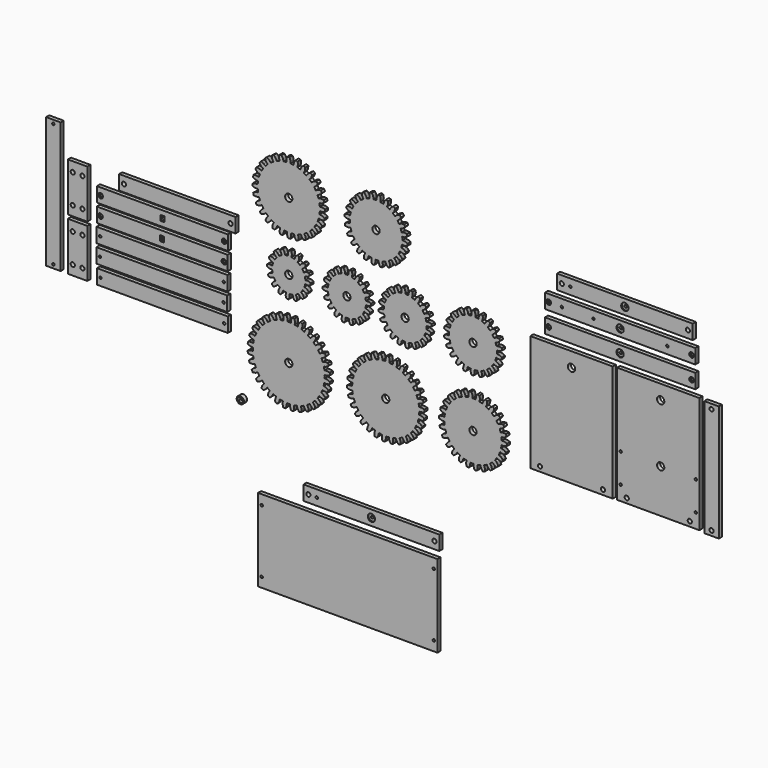
from build123d import *

# Parameters (mm, degrees)
F0_W      = 185.0000001032
F0_H      = 85
F0_R      = 1.25
F1_DEPTH  = 4
F0_W_2    = 140
F0_H_2    = 15
F0_R_2    = 2.15
F0_R_3    = 3.75
F2_DEPTH  = 3
F3_W      = 85
F3_H      = 120
F3_R      = 2.1499999403
F3_R_2    = 2.1500001135
F3_R_3    = 3.7499998228
F4_DEPTH  = 4
F3_R_4    = 1.2500001368
F3_R_5    = 1.2499999189
F3_R_6    = 2.1500001363
F3_R_7    = 3.7500003334
F3_R_8    = 2.1500001771
F3_R_9    = 1.2499998384
F3_R_10   = 1.2499998816
F3_R_11   = 3.7499998642
F3_W_2    = 15
F3_R_12   = 2.1499999772
F3_R_13   = 2.1499999639
F3_W_3    = 155
F3_H_2    = 15
F3_R_14   = 2.5000002092
F3_R_15   = 3.7500001582
F3_R_16   = 2.4999998652
F3_R_17   = 2.4999999715
F3_R_18   = 1.2500002315
F3_R_19   = 1.2499997471
F3_R_20   = 3.7500002135
F3_R_21   = 1.2499998097
F3_R_22   = 2.4999999683
F3_W_4    = 140
F3_R_23   = 2.1500001668
F3_R_24   = 1.2500002226
F3_R_25   = 3.7500004509
F3_R_26   = 2.1499998474
F3_R_27   = 1.2500000096
F5_DEPTH  = 3
F3_R_28   = 1.2500002694
F3_R_29   = 1.2500002977
F3_R_30   = 1.2500000055
F3_R_31   = 1.2500000442
F3_R_32   = 1.2499999628
F3_R_33   = 1.2500000631
F6_W      = 120
F6_H      = 15
F6_R      = 2.1499998407
F6_R_2    = 2.1500001203
F7_DEPTH  = 4
F6_W_2    = 135
F6_R_3    = 2.5000003053
F6_W_3    = 4.2
F6_H_2    = 5.5
F6_R_4    = 2.500000152
F6_R_5    = 2.4999997723
F6_R_6    = 2.4999998523
F6_R_7    = 1.2499997923
F6_R_8    = 1.2499998293
F6_R_9    = 1.24999975
F6_R_10   = 1.2500002277
F6_R_11   = 1.2500000547
F6_R_12   = 1.2500001786
F6_W_4    = 20
F6_H_3    = 50
F6_R_13   = 2.1499999167
F6_R_14   = 2.1500002553
F6_R_15   = 2.149999997
F6_R_16   = 2.1499998987
F6_W_5    = 15
F6_H_4    = 135
F6_R_17   = 1.249999987
F6_R_18   = 1.2499997585
F6_R_19   = 2.1500000538
F6_R_20   = 2.1500000872
F6_R_21   = 2.150000214
F6_R_22   = 2.1500000418
F6_R_23   = 1.2499995498
F6_R_24   = 1.2500001511
F6_R_25   = 1.2499999663
F8_DEPTH  = 3
F6_R_26   = 1.2499997721
F6_R_27   = 1.2499999151
F6_R_28   = 1.2499999183
F9_R      = 3.75
F9_W      = 6
F9_H      = 4.1362
F10_DEPTH = 4


# Not quite as in the source:
# - ends of sketch curves that miss each other by under 0.0002 mm in the source are joined


with BuildPart() as f1:
    # F0 (on Front) → F1 (new body)
    with BuildSketch(Plane.XZ):
        with Locations((-33.3591177641, -237.3350372048)):
            Rectangle(F0_W, F0_H)
        with Locations((-122.109118262, -269.8350372741)):
            Circle(F0_R, mode=Mode.SUBTRACT)
        with Locations((55.3908817492, -269.8350367553)):
            Circle(F0_R, mode=Mode.SUBTRACT)
        with Locations((-122.1091184837, -204.8350366392)):
            Circle(F0_R, mode=Mode.SUBTRACT)
        with Locations((55.390881907, -204.8350374057)):
            Circle(F0_R, mode=Mode.SUBTRACT)
    extrude(amount=F1_DEPTH)


with BuildPart() as f1b:
    # F0 (on Front) → F1, piece 2 (new body)
    with BuildSketch(Plane.XZ):
        with Locations((-8.9992198157, -179.4368852048)):
            Rectangle(F0_W_2, F0_H_2)
        with Locations((-73.9992204729, -179.43688553)):
            Circle(F0_R_2, mode=Mode.SUBTRACT)
        with Locations((-65.249220169, -179.4368847353)):
            Circle(F0_R, mode=Mode.SUBTRACT)
        with Locations((-8.9992199417, -179.4368858143)):
            Circle(F0_R_3, mode=Mode.SUBTRACT)
        with Locations((56.000779357, -179.43688553)):
            Circle(F0_R_2, mode=Mode.SUBTRACT)
    extrude(amount=F1_DEPTH)

    # F0 (on Front) → F2 (join)
    with BuildSketch(Plane.XZ):
        with Locations((-8.9992199417, -179.4368858143)):
            Circle(F0_R_3)
        with Locations((-8.9992199417, -179.4368858143)):
            Circle(F0_R, mode=Mode.SUBTRACT)
    extrude(amount=F2_DEPTH)


with BuildPart() as f4:
    # F3 (on Front) → F4 (new body)
    with BuildSketch(Plane.XZ):
        with Locations((197.3920837915, -21.156775845)):
            Rectangle(F3_W, F3_H)
        with Locations((164.8920831138, -76.1567756255)):
            Circle(F3_R, mode=Mode.SUBTRACT)
        with Locations((229.8920834124, -76.1567757998)):
            Circle(F3_R_2, mode=Mode.SUBTRACT)
        with Locations((197.3920835776, 23.8432242405)):
            Circle(F3_R_3, mode=Mode.SUBTRACT)
    extrude(amount=F4_DEPTH)


with BuildPart() as f4b:
    # F3 (on Front) → F4, piece 2 (new body)
    with BuildSketch(Plane.XZ):
        with Locations((286.8773457915, -20.760960845)):
            Rectangle(F3_W, F3_H)
        with Locations((248.1273454096, -65.7609605339)):
            Circle(F3_R_4, mode=Mode.SUBTRACT)
        with Locations((248.1273459001, -35.7609608013)):
            Circle(F3_R_5, mode=Mode.SUBTRACT)
        with Locations((254.3773459754, -75.7609612118)):
            Circle(F3_R_6, mode=Mode.SUBTRACT)
        with Locations((289.3773459928, -35.7609608746)):
            Circle(F3_R_7, mode=Mode.SUBTRACT)
        with Locations((319.3773460899, -75.7609608865)):
            Circle(F3_R_8, mode=Mode.SUBTRACT)
        with Locations((325.6273459002, -65.7609609473)):
            Circle(F3_R_9, mode=Mode.SUBTRACT)
        with Locations((325.6273463688, -35.7609615116)):
            Circle(F3_R_10, mode=Mode.SUBTRACT)
        with Locations((289.3773462437, 24.2390388005)):
            Circle(F3_R_11, mode=Mode.SUBTRACT)
    extrude(amount=F4_DEPTH)


with BuildPart() as f4c:
    # F3 (on Front) → F4, piece 3 (new body)
    with BuildSketch(Plane.XZ):
        with Locations((341.8244987915, -21.831593845)):
            Rectangle(F3_W_2, F3_H)
        with Locations((341.8244987664, -76.8315933296)):
            Circle(F3_R_12, mode=Mode.SUBTRACT)
        with Locations((341.8244990447, 33.1684061612)):
            Circle(F3_R_13, mode=Mode.SUBTRACT)
    extrude(amount=F4_DEPTH)


with BuildPart() as f4d:
    # F3 (on Front) → F4, piece 4 (new body)
    with BuildSketch(Plane.XZ):
        with Locations((247.5308627915, 53.263479155)):
            Rectangle(F3_W_3, F3_H_2)
        with Locations((173.780862357, 53.2634791719)):
            Circle(F3_R_14, mode=Mode.SUBTRACT)
        with Locations((247.530863227, 53.2634796235)):
            Circle(F3_R_15, mode=Mode.SUBTRACT)
        with Locations((321.2808632354, 53.2634795888)):
            Circle(F3_R_16, mode=Mode.SUBTRACT)
    extrude(amount=F4_DEPTH)

    # F3 (on Front) → F5, piece 3 (join)
    with BuildSketch(Plane.XZ):
        with Locations((247.530863227, 53.2634796235)):
            Circle(F3_R_15)
        with Locations((247.5308626029, 53.26347949)):
            Circle(F3_R_31, mode=Mode.SUBTRACT)
        with Locations((173.780862357, 53.2634791719)):
            Circle(F3_R_14)
        with Locations((173.7808627573, 53.2634792182)):
            Circle(F3_R_32, mode=Mode.SUBTRACT)
        with Locations((321.2808632354, 53.2634795888)):
            Circle(F3_R_16)
        with Locations((321.2808631303, 53.2634789986)):
            Circle(F3_R_33, mode=Mode.SUBTRACT)
    extrude(amount=F5_DEPTH)


with BuildPart() as f4e:
    # F3 (on Front) → F4, piece 5 (new body)
    with BuildSketch(Plane.XZ):
        with Locations((247.5308627915, 75.763479155)):
            Rectangle(F3_W_3, F3_H_2)
        with Locations((173.7808629702, 75.7634797471)):
            Circle(F3_R_17, mode=Mode.SUBTRACT)
        with Locations((187.5308632886, 75.7634786507)):
            Circle(F3_R_18, mode=Mode.SUBTRACT)
        with Locations((220.0308638283, 75.76347922)):
            Circle(F3_R_19, mode=Mode.SUBTRACT)
        with Locations((247.5308628153, 75.7634792893)):
            Circle(F3_R_20, mode=Mode.SUBTRACT)
        with Locations((296.2808628373, 75.7634789647)):
            Circle(F3_R_21, mode=Mode.SUBTRACT)
        with Locations((321.2808629677, 75.7634789591)):
            Circle(F3_R_22, mode=Mode.SUBTRACT)
    extrude(amount=F4_DEPTH)

    # F3 (on Front) → F5, piece 2 (join)
    with BuildSketch(Plane.XZ):
        with Locations((247.5308628153, 75.7634792893)):
            Circle(F3_R_20)
        with Locations((247.5308627907, 75.763479565)):
            Circle(F3_R_28, mode=Mode.SUBTRACT)
        with Locations((173.7808629702, 75.7634797471)):
            Circle(F3_R_17)
        with Locations((173.7808628831, 75.7634790697)):
            Circle(F3_R_29, mode=Mode.SUBTRACT)
        with Locations((321.2808629677, 75.7634789591)):
            Circle(F3_R_22)
        with Locations((321.2808631274, 75.7634793457)):
            Circle(F3_R_30, mode=Mode.SUBTRACT)
    extrude(amount=F5_DEPTH)


with BuildPart() as f4f:
    # F3 (on Front) → F4, piece 6 (new body)
    with BuildSketch(Plane.XZ):
        with Locations((252.3880877915, 97.053322155)):
            Rectangle(F3_W_4, F3_H_2)
        with Locations((187.3880875016, 97.0533224442)):
            Circle(F3_R_23, mode=Mode.SUBTRACT)
        with Locations((196.1380872713, 97.0533226464)):
            Circle(F3_R_24, mode=Mode.SUBTRACT)
        with Locations((252.3880869924, 97.0533221056)):
            Circle(F3_R_25, mode=Mode.SUBTRACT)
        with Locations((317.3880871466, 97.0533221238)):
            Circle(F3_R_26, mode=Mode.SUBTRACT)
    extrude(amount=F4_DEPTH)

    # F3 (on Front) → F5 (join)
    with BuildSketch(Plane.XZ):
        with Locations((252.3880869924, 97.0533221056)):
            Circle(F3_R_25)
        with Locations((252.3880872435, 97.0533220907)):
            Circle(F3_R_27, mode=Mode.SUBTRACT)
    extrude(amount=F5_DEPTH)


with BuildPart() as f7:
    # F6 (on Front) → F7 (new body)
    with BuildSketch(Plane.XZ):
        with Locations((-209.1869192228, 40.5194736201)):
            Rectangle(F6_W, F6_H)
        with Locations((-264.1869186715, 40.519473395)):
            Circle(F6_R, mode=Mode.SUBTRACT)
        with Locations((-154.1869191047, 40.5194738801)):
            Circle(F6_R_2, mode=Mode.SUBTRACT)
    extrude(amount=F7_DEPTH)


with BuildPart() as f7b:
    # F6 (on Front) → F7, piece 2 (new body)
    with BuildSketch(Plane.XZ):
        with Locations((-224.5559232228, 22.1369526201)):
            Rectangle(F6_W_2, F6_H)
        with Locations((-288.3059234909, 22.1369527791)):
            Circle(F6_R_3, mode=Mode.SUBTRACT)
        with Locations((-224.5559232228, 22.1369526201)):
            Rectangle(F6_W_3, F6_H_2, mode=Mode.SUBTRACT)
        with Locations((-160.8059236547, 22.1369530205)):
            Circle(F6_R_4, mode=Mode.SUBTRACT)
    extrude(amount=F7_DEPTH)

    # F6 (on Front) → F8 (join)
    with BuildSketch(Plane.XZ):
        with Locations((-288.3059234909, 22.1369527791)):
            Circle(F6_R_3)
        with Locations((-288.3059237228, 22.1369527941)):
            Circle(F6_R_23, mode=Mode.SUBTRACT)
        with Locations((-224.5559232228, 22.1369526201)):
            Rectangle(F6_W_3, F6_H_2)
        with Locations((-224.5559238074, 22.1369523654)):
            Circle(F6_R_24, mode=Mode.SUBTRACT)
        with Locations((-160.8059236547, 22.1369530205)):
            Circle(F6_R_4)
        with Locations((-160.8059232668, 22.1369526137)):
            Circle(F6_R_25, mode=Mode.SUBTRACT)
    extrude(amount=F8_DEPTH)


with BuildPart() as f7c:
    # F6 (on Front) → F7, piece 3 (new body)
    with BuildSketch(Plane.XZ):
        with Locations((-224.7267092228, 3.5650316201)):
            Rectangle(F6_W_2, F6_H)
        with Locations((-288.4767094247, 3.5650314574)):
            Circle(F6_R_5, mode=Mode.SUBTRACT)
        with Locations((-224.7267092228, 3.5650316201)):
            Rectangle(F6_W_3, F6_H_2, mode=Mode.SUBTRACT)
        with Locations((-160.9767097593, 3.5650311037)):
            Circle(F6_R_6, mode=Mode.SUBTRACT)
    extrude(amount=F7_DEPTH)

    # F6 (on Front) → F8, piece 2 (join)
    with BuildSketch(Plane.XZ):
        with Locations((-288.4767094247, 3.5650314574)):
            Circle(F6_R_5)
        with Locations((-288.4767097646, 3.5650314288)):
            Circle(F6_R_26, mode=Mode.SUBTRACT)
        with Locations((-224.7267092228, 3.5650316201)):
            Rectangle(F6_W_3, F6_H_2)
        with Locations((-224.7267099234, 3.5650315072)):
            Circle(F6_R_27, mode=Mode.SUBTRACT)
        with Locations((-160.9767097593, 3.5650311037)):
            Circle(F6_R_6)
        with Locations((-160.9767096346, 3.5650313951)):
            Circle(F6_R_28, mode=Mode.SUBTRACT)
    extrude(amount=F8_DEPTH)


with BuildPart() as f7d:
    # F6 (on Front) → F7, piece 4 (new body)
    with BuildSketch(Plane.XZ):
        with Locations((-224.9429642228, -14.8729813799)):
            Rectangle(F6_W_2, F6_H)
        with Locations((-288.6929639963, -14.8729814839)):
            Circle(F6_R_7, mode=Mode.SUBTRACT)
        with Locations((-161.1929638922, -14.872981641)):
            Circle(F6_R_8, mode=Mode.SUBTRACT)
    extrude(amount=F7_DEPTH)


with BuildPart() as f7e:
    # F6 (on Front) → F7, piece 5 (new body)
    with BuildSketch(Plane.XZ):
        with Locations((-225.2052152228, -33.4813383799)):
            Rectangle(F6_W_2, F6_H)
        with Locations((-288.9552157179, -33.4813383275)):
            Circle(F6_R_9, mode=Mode.SUBTRACT)
        with Locations((-161.455215521, -33.4813382143)):
            Circle(F6_R_10, mode=Mode.SUBTRACT)
    extrude(amount=F7_DEPTH)


with BuildPart() as f7f:
    # F6 (on Front) → F7, piece 6 (new body)
    with BuildSketch(Plane.XZ):
        with Locations((-224.6013922228, -52.3583963799)):
            Rectangle(F6_W_2, F6_H)
        with Locations((-288.3513919109, -52.3583972026)):
            Circle(F6_R_11, mode=Mode.SUBTRACT)
        with Locations((-160.8513918034, -52.3583971174)):
            Circle(F6_R_12, mode=Mode.SUBTRACT)
    extrude(amount=F7_DEPTH)


with BuildPart() as f7g:
    # F6 (on Front) → F7, piece 7 (new body)
    with BuildSketch(Plane.XZ):
        with Locations((-311.9977712228, -34.7509243799)):
            Rectangle(F6_W_4, F6_H_3)
        with Locations((-316.9977711889, -49.7509249127)):
            Circle(F6_R_13, mode=Mode.SUBTRACT)
        with Locations((-306.9977711289, -49.7509244579)):
            Circle(F6_R_14, mode=Mode.SUBTRACT)
        with Locations((-316.9977717293, -19.7509244938)):
            Circle(F6_R_15, mode=Mode.SUBTRACT)
        with Locations((-306.9977710666, -19.750924159)):
            Circle(F6_R_16, mode=Mode.SUBTRACT)
    extrude(amount=F7_DEPTH)


with BuildPart() as f7h:
    # F6 (on Front) → F7, piece 8 (new body)
    with BuildSketch(Plane.XZ):
        with Locations((-336.9977712228, 7.7490756201)):
            Rectangle(F6_W_5, F6_H_4)
        with Locations((-336.9977717711, -56.000924598)):
            Circle(F6_R_17, mode=Mode.SUBTRACT)
        with Locations((-336.9977713756, 71.4990756451)):
            Circle(F6_R_18, mode=Mode.SUBTRACT)
    extrude(amount=F7_DEPTH)


with BuildPart() as f7i:
    # F6 (on Front) → F7, piece 9 (new body)
    with BuildSketch(Plane.XZ):
        with Locations((-311.9977712228, 19.1153636201)):
            Rectangle(F6_W_4, F6_H_3)
        with Locations((-316.997771029, 4.1153636536)):
            Circle(F6_R_19, mode=Mode.SUBTRACT)
        with Locations((-306.9977714868, 4.1153634701)):
            Circle(F6_R_20, mode=Mode.SUBTRACT)
        with Locations((-316.9977715309, 34.1153632565)):
            Circle(F6_R_21, mode=Mode.SUBTRACT)
        with Locations((-306.9977714155, 34.1153636931)):
            Circle(F6_R_22, mode=Mode.SUBTRACT)
    extrude(amount=F7_DEPTH)


with BuildPart() as f10:
    # F9 (on Front) → F10 (new body)
    with BuildSketch(Plane.XZ):
        with Locations((-144.19643, -116.58612)):
            Circle(F9_R)
        with Locations((-144.19643, -116.58612)):
            Rectangle(F9_W, F9_H, mode=Mode.SUBTRACT)
    extrude(amount=F10_DEPTH)


with BuildPart() as f10b:
    # F9 (on Front) → F10, piece 2 (new body)
    with BuildSketch(Plane.XZ):
        with BuildLine():
            Line((-65.34288, -40.75651), (-66.54871, -41.83597))
            ThreePointArc((-66.54871, -41.83597), (-67.6510340915, -40.6572073288), (-68.8035722148, -39.5274923601))
            Line((-68.8035722148, -39.5274923601), (-67.69609, -38.34736))
            Line((-67.69609, -38.34736), (-67.66416, -38.31098))
            Line((-67.66416, -38.31098), (-67.57332, -38.19769))
            Line((-67.57332, -38.19769), (-67.43133, -38.00171))
            Line((-67.43133, -38.00171), (-67.24638, -37.71783))
            Line((-67.24638, -37.71783), (-67.02701, -37.34147))
            Line((-67.02701, -37.34147), (-66.78214, -36.8687))
            Line((-66.78214, -36.8687), (-66.52097, -36.29623))
            Line((-66.52097, -36.29623), (-66.25296, -35.62147))
            Line((-66.25296, -35.62147), (-65.98775, -34.84254))
            Line((-65.98775, -34.84254), (-65.97748, -34.80656))
            ThreePointArc((-65.97748, -34.80656), (-66.8506396677, -34.0521723283), (-67.7439610985, -33.3217713814))
            Line((-67.7439610985, -33.3217713814), (-67.77764, -33.33809))
            Line((-67.77764, -33.33809), (-68.49935, -33.73331))
            Line((-68.49935, -33.73331), (-69.11795, -34.11339))
            Line((-69.11795, -34.11339), (-69.63697, -34.46912))
            Line((-69.63697, -34.46912), (-70.06059, -34.79166))
            Line((-70.06059, -34.79166), (-70.39361, -35.07249))
            Line((-70.39361, -35.07249), (-70.64144, -35.30351))
            Line((-70.64144, -35.30351), (-70.81008, -35.4771))
            Line((-70.81008, -35.4771), (-70.90605, -35.58606))
            Line((-70.90605, -35.58606), (-70.9364, -35.62377))
            Line((-70.9364, -35.62377), (-71.90847, -36.91773))
            ThreePointArc((-71.90847, -36.91773), (-73.2195810441, -35.9766710646), (-74.5703711366, -35.0935118238))
            Line((-74.5703711366, -35.0935118238), (-73.7144, -33.72))
            Line((-73.7144, -33.72), (-73.69018, -33.67809))
            Line((-73.69018, -33.67809), (-73.62319, -33.54926))
            Line((-73.62319, -33.54926), (-73.52216, -33.32934))
            Line((-73.52216, -33.32934), (-73.39614, -33.01483))
            Line((-73.39614, -33.01483), (-73.25441, -32.60291))
            Line((-73.25441, -32.60291), (-73.10648, -32.09145))
            Line((-73.10648, -32.09145), (-72.96201, -31.47903))
            Line((-72.96201, -31.47903), (-72.83079, -30.76495))
            Line((-72.83079, -30.76495), (-72.72264, -29.94925))
            Line((-72.72264, -29.94925), (-72.71958, -29.91195))
            ThreePointArc((-72.71958, -29.91195), (-73.7231375628, -29.3424051372), (-74.7417883799, -28.8003168534))
            Line((-74.7417883799, -28.8003168534), (-74.77164, -28.82289))
            Line((-74.77164, -28.82289), (-75.40238, -29.35131))
            Line((-75.40238, -29.35131), (-75.93495, -29.84477))
            Line((-75.93495, -29.84477), (-76.37459, -30.29493))
            Line((-76.37459, -30.29493), (-76.72714, -30.69391))
            Line((-76.72714, -30.69391), (-76.99898, -31.03431))
            Line((-76.99898, -31.03431), (-77.19698, -31.30925))
            Line((-77.19698, -31.30925), (-77.32851, -31.5124))
            Line((-77.32851, -31.5124), (-77.40138, -31.638))
            Line((-77.40138, -31.638), (-77.42379, -31.6809))
            Line((-77.42379, -31.6809), (-78.12474, -33.13963))
            ThreePointArc((-78.12474, -33.13963), (-79.5942507744, -32.4724435914), (-81.091380201, -31.8697805326))
            Line((-81.091380201, -31.8697805326), (-80.51982, -30.35566))
            Line((-80.51982, -30.35566), (-80.50424, -30.30983))
            Line((-80.50424, -30.30983), (-80.46367, -30.17041))
            Line((-80.46367, -30.17041), (-80.40749, -29.93501))
            Line((-80.40749, -29.93501), (-80.34524, -29.60196))
            Line((-80.34524, -29.60196), (-80.2866, -29.1703))
            Line((-80.2866, -29.1703), (-80.2413, -28.63981))
            Line((-80.2413, -28.63981), (-80.21908, -28.01097))
            Line((-80.21908, -28.01097), (-80.22969, -27.28501))
            Line((-80.22969, -27.28501), (-80.28275, -26.46388))
            Line((-80.28275, -26.46388), (-80.28703, -26.42671))
            ThreePointArc((-80.28703, -26.42671), (-81.3824159287, -26.0638909969), (-82.4872493906, -25.7309478738))
            Line((-82.4872493906, -25.7309478738), (-82.51212, -25.75891))
            Line((-82.51212, -25.75891), (-83.02765, -26.40023))
            Line((-83.02765, -26.40023), (-83.45372, -26.98811))
            Line((-83.45372, -26.98811), (-83.79709, -27.51539))
            Line((-83.79709, -27.51539), (-84.06503, -27.97548))
            Line((-84.06503, -27.97548), (-84.26523, -28.36237))
            Line((-84.26523, -28.36237), (-84.40579, -28.67066))
            Line((-84.40579, -28.67066), (-84.49517, -28.89556))
            Line((-84.49517, -28.89556), (-84.54214, -29.03296))
            Line((-84.54214, -29.03296), (-84.55574, -29.07942))
            Line((-84.55574, -29.07942), (-84.95864, -30.64687))
            ThreePointArc((-84.95864, -30.64687), (-86.5300739656, -30.2791848305), (-88.1160095461, -29.9801772672))
            Line((-88.1160095461, -29.9801772672), (-87.85082, -28.38365))
            Line((-87.85082, -28.38365), (-87.84448, -28.33566))
            Line((-87.84448, -28.33566), (-87.83189, -28.191))
            Line((-87.83189, -28.191), (-87.82271, -27.94916))
            Line((-87.82271, -27.94916), (-87.82664, -27.61037))
            Line((-87.82664, -27.61037), (-87.85334, -27.17556))
            Line((-87.85334, -27.17556), (-87.9124, -26.64642))
            Line((-87.9124, -26.64642), (-88.01329, -26.02533))
            Line((-88.01329, -26.02533), (-88.16532, -25.31539))
            Line((-88.16532, -25.31539), (-88.37756, -24.5204))
            Line((-88.37756, -24.5204), (-88.38901, -24.48477))
            ThreePointArc((-88.38901, -24.48477), (-89.53413141, -24.3426237922), (-90.682690038, -24.2316204577))
            Line((-90.682690038, -24.2316204577), (-90.70163, -24.2639))
            Line((-90.70163, -24.2639), (-91.08213, -24.99347))
            Line((-91.08213, -24.99347), (-91.38532, -25.65317))
            Line((-91.38532, -25.65317), (-91.61923, -26.23731))
            Line((-91.61923, -26.23731), (-91.79227, -26.74083))
            Line((-91.79227, -26.74083), (-91.91314, -27.15935))
            Line((-91.91314, -27.15935), (-91.99086, -27.48913))
            Line((-91.99086, -27.48913), (-92.03464, -27.72715))
            Line((-92.03464, -27.72715), (-92.0539, -27.87108))
            Line((-92.0539, -27.87108), (-92.05818, -27.91929))
            Line((-92.05818, -27.91929), (-92.14754, -29.53523))
            ThreePointArc((-92.14754, -29.53523), (-93.7605126768, -29.4811805399), (-95.3743100297, -29.4973190638))
            Line((-95.3743100297, -29.4973190638), (-95.42568, -27.87973))
            Line((-95.42568, -27.87973), (-95.42883, -27.83143))
            Line((-95.42883, -27.83143), (-95.4447, -27.68709))
            Line((-95.4447, -27.68709), (-95.48288, -27.44811))
            Line((-95.48288, -27.44811), (-95.55283, -27.11659))
            Line((-95.55283, -27.11659), (-95.66384, -26.69535))
            Line((-95.66384, -26.69535), (-95.82499, -26.1879))
            Line((-95.82499, -26.1879), (-96.04512, -25.59843))
            Line((-96.04512, -25.59843), (-96.33272, -24.93179))
            Line((-96.33272, -24.93179), (-96.69598, -24.19347))
            Line((-96.69598, -24.19347), (-96.71416, -24.16076))
            ThreePointArc((-96.71416, -24.16076), (-97.8650119246, -24.2447512613), (-99.0131595723, -24.3599537494))
            Line((-99.0131595723, -24.3599537494), (-99.02544, -24.39531))
            Line((-99.02544, -24.39531), (-99.2563, -25.1851))
            Line((-99.2563, -25.1851), (-99.42496, -25.89127))
            Line((-99.42496, -25.89127), (-99.54042, -26.50982))
            Line((-99.54042, -26.50982), (-99.61189, -27.03742))
            Line((-99.61189, -27.03742), (-99.6488, -27.47148))
            Line((-99.6488, -27.47148), (-99.66068, -27.81009))
            Line((-99.66068, -27.81009), (-99.65719, -28.05207))
            Line((-99.65719, -28.05207), (-99.648, -28.19699))
            Line((-99.648, -28.19699), (-99.64279, -28.24511))
            Line((-99.64279, -28.24511), (-99.41518, -29.84743))
            ThreePointArc((-99.41518, -29.84743), (-101.0077015469, -30.1090979702), (-102.5873395258, -30.4397620427))
            Line((-102.5873395258, -30.4397620427), (-102.9533, -28.86328))
            Line((-102.9533, -28.86328), (-102.96582, -28.81652))
            Line((-102.96582, -28.81652), (-103.00954, -28.67805))
            Line((-103.00954, -28.67805), (-103.09361, -28.45111))
            Line((-103.09361, -28.45111), (-103.22689, -28.13961))
            Line((-103.22689, -28.13961), (-103.41794, -27.74812))
            Line((-103.41794, -27.74812), (-103.675, -27.28186))
            Line((-103.675, -27.28186), (-104.0059, -26.74666))
            Line((-104.0059, -26.74666), (-104.41803, -26.14893))
            Line((-104.41803, -26.14893), (-104.91835, -25.49568))
            Line((-104.91835, -25.49568), (-104.94256, -25.46714))
            ThreePointArc((-104.94256, -25.46714), (-106.0549105461, -25.7740330755), (-107.1585188996, -26.1110134361))
            Line((-107.1585188996, -26.1110134361), (-107.16367, -26.14808))
            Line((-107.16367, -26.14808), (-107.23601, -26.96774))
            Line((-107.23601, -26.96774), (-107.26367, -27.69324))
            Line((-107.26367, -27.69324), (-107.25623, -28.32243))
            Line((-107.25623, -28.32243), (-107.2234, -28.85384))
            Line((-107.2234, -28.85384), (-107.17492, -29.28676))
            Line((-107.17492, -29.28676), (-107.12052, -29.62118))
            Line((-107.12052, -29.62118), (-107.06988, -29.85783))
            Line((-107.06988, -29.85783), (-107.03259, -29.99817))
            Line((-107.03259, -29.99817), (-107.0181, -30.04436))
            Line((-107.0181, -30.04436), (-106.48227, -31.57148))
            ThreePointArc((-106.48227, -31.57148), (-107.9931425453, -32.1388083605), (-109.4779193991, -32.7712913298))
            Line((-109.4779193991, -32.7712913298), (-110.14441, -31.29649))
            Line((-110.14441, -31.29649), (-110.1658, -31.25307))
            Line((-110.1658, -31.25307), (-110.2357, -31.1258))
            Line((-110.2357, -31.1258), (-110.36242, -30.91962))
            Line((-110.36242, -30.91962), (-110.55391, -30.6401))
            Line((-110.55391, -30.6401), (-110.81767, -30.29341))
            Line((-110.81767, -30.29341), (-111.16075, -29.88626))
            Line((-111.16075, -29.88626), (-111.5897, -29.42589))
            Line((-111.5897, -29.42589), (-112.11053, -28.92006))
            Line((-112.11053, -28.92006), (-112.72868, -28.37696))
            Line((-112.72868, -28.37696), (-112.75799, -28.35369))
            ThreePointArc((-112.75799, -28.35369), (-113.7890958692, -28.8717004215), (-114.8057597012, -29.4175105389))
            Line((-114.8057597012, -29.4175105389), (-114.80358, -29.45487))
            Line((-114.80358, -29.45487), (-114.71462, -30.27289))
            Line((-114.71462, -30.27289), (-114.60021, -30.98985))
            Line((-114.60021, -30.98985), (-114.47017, -31.6055))
            Line((-114.47017, -31.6055), (-114.3343, -32.12029))
            Line((-114.3343, -32.12029), (-114.20229, -32.53543))
            Line((-114.20229, -32.53543), (-114.08369, -32.85281))
            Line((-114.08369, -32.85281), (-113.98785, -33.07504))
            Line((-113.98785, -33.07504), (-113.92391, -33.20541))
            Line((-113.92391, -33.20541), (-113.90068, -33.24788))
            Line((-113.90068, -33.24788), (-113.07721, -34.64113))
            ThreePointArc((-113.07721, -34.64113), (-114.4483781204, -35.4923078571), (-115.7812364238, -36.4023050009))
            Line((-115.7812364238, -36.4023050009), (-116.72263, -35.08587))
            Line((-116.72263, -35.08587), (-116.75209, -35.04746))
            Line((-116.75209, -35.04746), (-116.84547, -34.93626))
            Line((-116.84547, -34.93626), (-117.00999, -34.75877))
            Line((-117.00999, -34.75877), (-117.25233, -34.52198))
            Line((-117.25233, -34.52198), (-117.57866, -34.23341))
            Line((-117.57866, -34.23341), (-117.99458, -33.90101))
            Line((-117.99458, -33.90101), (-118.5051, -33.53317))
            Line((-118.5051, -33.53317), (-119.1146, -33.13867))
            Line((-119.1146, -33.13867), (-119.82682, -32.7266))
            Line((-119.82682, -32.7266), (-119.86011, -32.7095))
            ThreePointArc((-119.86011, -32.7095), (-120.7703444706, -33.4187102472), (-121.6609885171, -34.1523717513))
            Line((-121.6609885171, -34.1523717513), (-121.65156, -34.18859))
            Line((-121.65156, -34.18859), (-121.40473, -34.97354))
            Line((-121.40473, -34.97354), (-121.15264, -35.6544))
            Line((-121.15264, -35.6544), (-120.90499, -36.23285))
            Line((-120.90499, -36.23285), (-120.6713, -36.71125))
            Line((-120.6713, -36.71125), (-120.46084, -37.09266))
            Line((-120.46084, -37.09266), (-120.2826, -37.3808))
            Line((-120.2826, -37.3808), (-120.14525, -37.58006))
            Line((-120.14525, -37.58006), (-120.0571, -37.69545))
            Line((-120.0571, -37.69545), (-120.02604, -37.73257))
            Line((-120.02604, -37.73257), (-118.94658, -38.9384))
            ThreePointArc((-118.94658, -38.9384), (-120.1253426712, -40.0407240915), (-121.2550576399, -41.1932622148))
            Line((-121.2550576399, -41.1932622148), (-122.43519, -40.08578))
            Line((-122.43519, -40.08578), (-122.47157, -40.05385))
            Line((-122.47157, -40.05385), (-122.58486, -39.96301))
            Line((-122.58486, -39.96301), (-122.78084, -39.82102))
            Line((-122.78084, -39.82102), (-123.06472, -39.63607))
            Line((-123.06472, -39.63607), (-123.44108, -39.4167))
            Line((-123.44108, -39.4167), (-123.91385, -39.17183))
            Line((-123.91385, -39.17183), (-124.48632, -38.91066))
            Line((-124.48632, -38.91066), (-125.16108, -38.64265))
            Line((-125.16108, -38.64265), (-125.94001, -38.37744))
            Line((-125.94001, -38.37744), (-125.97599, -38.36717))
            ThreePointArc((-125.97599, -38.36717), (-126.7303776717, -39.2403296677), (-127.4607786186, -40.1336510985))
            Line((-127.4607786186, -40.1336510985), (-127.44446, -40.16733))
            Line((-127.44446, -40.16733), (-127.04924, -40.88904))
            Line((-127.04924, -40.88904), (-126.66916, -41.50764))
            Line((-126.66916, -41.50764), (-126.31343, -42.02666))
            Line((-126.31343, -42.02666), (-125.99089, -42.45028))
            Line((-125.99089, -42.45028), (-125.71006, -42.7833))
            Line((-125.71006, -42.7833), (-125.47904, -43.03113))
            Line((-125.47904, -43.03113), (-125.30545, -43.19977))
            Line((-125.30545, -43.19977), (-125.19649, -43.29574))
            Line((-125.19649, -43.29574), (-125.15878, -43.32609))
            Line((-125.15878, -43.32609), (-123.86482, -44.29816))
            ThreePointArc((-123.86482, -44.29816), (-124.8058789354, -45.6092710441), (-125.6890381762, -46.9600611366))
            Line((-125.6890381762, -46.9600611366), (-127.06255, -46.10409))
            Line((-127.06255, -46.10409), (-127.10446, -46.07987))
            Line((-127.10446, -46.07987), (-127.23329, -46.01288))
            Line((-127.23329, -46.01288), (-127.45321, -45.91185))
            Line((-127.45321, -45.91185), (-127.76772, -45.78583))
            Line((-127.76772, -45.78583), (-128.17964, -45.6441))
            Line((-128.17964, -45.6441), (-128.6911, -45.49617))
            Line((-128.6911, -45.49617), (-129.30352, -45.3517))
            Line((-129.30352, -45.3517), (-130.0176, -45.22048))
            Line((-130.0176, -45.22048), (-130.8333, -45.11233))
            Line((-130.8333, -45.11233), (-130.8706, -45.10927))
            ThreePointArc((-130.8706, -45.10927), (-131.4401448628, -46.1128275628), (-131.9822331466, -47.1314783799))
            Line((-131.9822331466, -47.1314783799), (-131.95966, -47.16133))
            Line((-131.95966, -47.16133), (-131.43124, -47.79207))
            Line((-131.43124, -47.79207), (-130.93778, -48.32464))
            Line((-130.93778, -48.32464), (-130.48762, -48.76428))
            Line((-130.48762, -48.76428), (-130.08864, -49.11683))
            Line((-130.08864, -49.11683), (-129.74824, -49.38867))
            Line((-129.74824, -49.38867), (-129.4733, -49.58667))
            Line((-129.4733, -49.58667), (-129.27015, -49.7182))
            Line((-129.27015, -49.7182), (-129.14455, -49.79107))
            Line((-129.14455, -49.79107), (-129.10165, -49.81348))
            Line((-129.10165, -49.81348), (-127.64292, -50.51443))
            ThreePointArc((-127.64292, -50.51443), (-128.3101064086, -51.9839407744), (-128.9127694674, -53.481070201))
            Line((-128.9127694674, -53.481070201), (-130.42689, -52.90951))
            Line((-130.42689, -52.90951), (-130.47272, -52.89393))
            Line((-130.47272, -52.89393), (-130.61214, -52.85336))
            Line((-130.61214, -52.85336), (-130.84754, -52.79718))
            Line((-130.84754, -52.79718), (-131.18059, -52.73493))
            Line((-131.18059, -52.73493), (-131.61225, -52.67629))
            Line((-131.61225, -52.67629), (-132.14274, -52.63099))
            Line((-132.14274, -52.63099), (-132.77158, -52.60877))
            Line((-132.77158, -52.60877), (-133.49754, -52.61938))
            Line((-133.49754, -52.61938), (-134.31867, -52.67244))
            Line((-134.31867, -52.67244), (-134.35584, -52.67672))
            ThreePointArc((-134.35584, -52.67672), (-134.7186590031, -53.7721059287), (-135.0516021262, -54.8769393906))
            Line((-135.0516021262, -54.8769393906), (-135.02364, -54.90181))
            Line((-135.02364, -54.90181), (-134.38232, -55.41734))
            Line((-134.38232, -55.41734), (-133.79444, -55.84341))
            Line((-133.79444, -55.84341), (-133.26716, -56.18678))
            Line((-133.26716, -56.18678), (-132.80707, -56.45472))
            Line((-132.80707, -56.45472), (-132.42018, -56.65492))
            Line((-132.42018, -56.65492), (-132.11189, -56.79548))
            Line((-132.11189, -56.79548), (-131.88699, -56.88486))
            Line((-131.88699, -56.88486), (-131.74959, -56.93183))
            Line((-131.74959, -56.93183), (-131.70313, -56.94543))
            Line((-131.70313, -56.94543), (-130.13568, -57.34833))
            ThreePointArc((-130.13568, -57.34833), (-130.5033651695, -58.9197639656), (-130.8023727328, -60.5056995461))
            Line((-130.8023727328, -60.5056995461), (-132.3989, -60.24051))
            Line((-132.3989, -60.24051), (-132.44689, -60.23417))
            Line((-132.44689, -60.23417), (-132.59155, -60.22158))
            Line((-132.59155, -60.22158), (-132.83339, -60.2124))
            Line((-132.83339, -60.2124), (-133.17218, -60.21633))
            Line((-133.17218, -60.21633), (-133.60699, -60.24303))
            Line((-133.60699, -60.24303), (-134.13613, -60.30209))
            Line((-134.13613, -60.30209), (-134.75722, -60.40298))
            Line((-134.75722, -60.40298), (-135.46716, -60.55501))
            Line((-135.46716, -60.55501), (-136.26215, -60.76725))
            Line((-136.26215, -60.76725), (-136.29778, -60.7787))
            ThreePointArc((-136.29778, -60.7787), (-136.4399262078, -61.92382141), (-136.5509295423, -63.072380038))
            Line((-136.5509295423, -63.072380038), (-136.51865, -63.09132))
            Line((-136.51865, -63.09132), (-135.78908, -63.47182))
            Line((-135.78908, -63.47182), (-135.12938, -63.77501))
            Line((-135.12938, -63.77501), (-134.54524, -64.00892))
            Line((-134.54524, -64.00892), (-134.04172, -64.18196))
            Line((-134.04172, -64.18196), (-133.6232, -64.30283))
            Line((-133.6232, -64.30283), (-133.29342, -64.38055))
            Line((-133.29342, -64.38055), (-133.0554, -64.42433))
            Line((-133.0554, -64.42433), (-132.91147, -64.44359))
            Line((-132.91147, -64.44359), (-132.86326, -64.44787))
            Line((-132.86326, -64.44787), (-131.24732, -64.53723))
            ThreePointArc((-131.24732, -64.53723), (-131.3013694601, -66.1502026768), (-131.2852309362, -67.7640000297))
            Line((-131.2852309362, -67.7640000297), (-132.90282, -67.81537))
            Line((-132.90282, -67.81537), (-132.95112, -67.81852))
            Line((-132.95112, -67.81852), (-133.09546, -67.83439))
            Line((-133.09546, -67.83439), (-133.33444, -67.87257))
            Line((-133.33444, -67.87257), (-133.66596, -67.94252))
            Line((-133.66596, -67.94252), (-134.0872, -68.05353))
            Line((-134.0872, -68.05353), (-134.59465, -68.21468))
            Line((-134.59465, -68.21468), (-135.18412, -68.43481))
            Line((-135.18412, -68.43481), (-135.85076, -68.72241))
            Line((-135.85076, -68.72241), (-136.58908, -69.08567))
            Line((-136.58908, -69.08567), (-136.62179, -69.10385))
            ThreePointArc((-136.62179, -69.10385), (-136.5377987387, -70.2547019246), (-136.4225962506, -71.4028495723))
            Line((-136.4225962506, -71.4028495723), (-136.38724, -71.41513))
            Line((-136.38724, -71.41513), (-135.59745, -71.64599))
            Line((-135.59745, -71.64599), (-134.89128, -71.81465))
            Line((-134.89128, -71.81465), (-134.27273, -71.93011))
            Line((-134.27273, -71.93011), (-133.74513, -72.00158))
            Line((-133.74513, -72.00158), (-133.31107, -72.03849))
            Line((-133.31107, -72.03849), (-132.97246, -72.05037))
            Line((-132.97246, -72.05037), (-132.73048, -72.04688))
            Line((-132.73048, -72.04688), (-132.58556, -72.03769))
            Line((-132.58556, -72.03769), (-132.53744, -72.03248))
            Line((-132.53744, -72.03248), (-130.93512, -71.80487))
            ThreePointArc((-130.93512, -71.80487), (-130.6734520298, -73.3973915469), (-130.3427879573, -74.9770295258))
            Line((-130.3427879573, -74.9770295258), (-131.91927, -75.34299))
            Line((-131.91927, -75.34299), (-131.96603, -75.35551))
            Line((-131.96603, -75.35551), (-132.1045, -75.39923))
            Line((-132.1045, -75.39923), (-132.33144, -75.4833))
            Line((-132.33144, -75.4833), (-132.64294, -75.61658))
            Line((-132.64294, -75.61658), (-133.03443, -75.80763))
            Line((-133.03443, -75.80763), (-133.50069, -76.06469))
            Line((-133.50069, -76.06469), (-134.03589, -76.39559))
            Line((-134.03589, -76.39559), (-134.63362, -76.80772))
            Line((-134.63362, -76.80772), (-135.28687, -77.30804))
            Line((-135.28687, -77.30804), (-135.31541, -77.33225))
            ThreePointArc((-135.31541, -77.33225), (-135.0085169245, -78.4446005461), (-134.6715365639, -79.5482088996))
            Line((-134.6715365639, -79.5482088996), (-134.63447, -79.55336))
            Line((-134.63447, -79.55336), (-133.81481, -79.6257))
            Line((-133.81481, -79.6257), (-133.08931, -79.65336))
            Line((-133.08931, -79.65336), (-132.46012, -79.64592))
            Line((-132.46012, -79.64592), (-131.92871, -79.61309))
            Line((-131.92871, -79.61309), (-131.49579, -79.56461))
            Line((-131.49579, -79.56461), (-131.16137, -79.51021))
            Line((-131.16137, -79.51021), (-130.92472, -79.45957))
            Line((-130.92472, -79.45957), (-130.78438, -79.42228))
            Line((-130.78438, -79.42228), (-130.73819, -79.40779))
            Line((-130.73819, -79.40779), (-129.21107, -78.87196))
            ThreePointArc((-129.21107, -78.87196), (-128.6437416395, -80.3828325453), (-128.0112586702, -81.8676093991))
            Line((-128.0112586702, -81.8676093991), (-129.48606, -82.5341))
            Line((-129.48606, -82.5341), (-129.52948, -82.55549))
            Line((-129.52948, -82.55549), (-129.65675, -82.62539))
            Line((-129.65675, -82.62539), (-129.86293, -82.75211))
            Line((-129.86293, -82.75211), (-130.14245, -82.9436))
            Line((-130.14245, -82.9436), (-130.48914, -83.20736))
            Line((-130.48914, -83.20736), (-130.89629, -83.55044))
            Line((-130.89629, -83.55044), (-131.35666, -83.97939))
            Line((-131.35666, -83.97939), (-131.86249, -84.50022))
            Line((-131.86249, -84.50022), (-132.40559, -85.11837))
            Line((-132.40559, -85.11837), (-132.42886, -85.14768))
            ThreePointArc((-132.42886, -85.14768), (-131.9108495785, -86.1787858692), (-131.3650394611, -87.1954497012))
            Line((-131.3650394611, -87.1954497012), (-131.32768, -87.19327))
            Line((-131.32768, -87.19327), (-130.50966, -87.10431))
            Line((-130.50966, -87.10431), (-129.7927, -86.9899))
            Line((-129.7927, -86.9899), (-129.17705, -86.85986))
            Line((-129.17705, -86.85986), (-128.66226, -86.72399))
            Line((-128.66226, -86.72399), (-128.24712, -86.59198))
            Line((-128.24712, -86.59198), (-127.92974, -86.47338))
            Line((-127.92974, -86.47338), (-127.70751, -86.37754))
            Line((-127.70751, -86.37754), (-127.57714, -86.3136))
            Line((-127.57714, -86.3136), (-127.53467, -86.29037))
            Line((-127.53467, -86.29037), (-126.14142, -85.4669))
            ThreePointArc((-126.14142, -85.4669), (-125.2902421429, -86.8380681204), (-124.3802449991, -88.1709264238))
            Line((-124.3802449991, -88.1709264238), (-125.69668, -89.11232))
            Line((-125.69668, -89.11232), (-125.73509, -89.14178))
            Line((-125.73509, -89.14178), (-125.84629, -89.23516))
            Line((-125.84629, -89.23516), (-126.02378, -89.39968))
            Line((-126.02378, -89.39968), (-126.26057, -89.64202))
            Line((-126.26057, -89.64202), (-126.54914, -89.96835))
            Line((-126.54914, -89.96835), (-126.88154, -90.38427))
            Line((-126.88154, -90.38427), (-127.24938, -90.89479))
            Line((-127.24938, -90.89479), (-127.64388, -91.50429))
            Line((-127.64388, -91.50429), (-128.05595, -92.21651))
            Line((-128.05595, -92.21651), (-128.07305, -92.2498))
            ThreePointArc((-128.07305, -92.2498), (-127.3638397528, -93.1600344706), (-126.6301782487, -94.0506785171))
            Line((-126.6301782487, -94.0506785171), (-126.59396, -94.04125))
            Line((-126.59396, -94.04125), (-125.80901, -93.79442))
            Line((-125.80901, -93.79442), (-125.12815, -93.54233))
            Line((-125.12815, -93.54233), (-124.5497, -93.29468))
            Line((-124.5497, -93.29468), (-124.0713, -93.06099))
            Line((-124.0713, -93.06099), (-123.68989, -92.85053))
            Line((-123.68989, -92.85053), (-123.40175, -92.67229))
            Line((-123.40175, -92.67229), (-123.20249, -92.53494))
            Line((-123.20249, -92.53494), (-123.0871, -92.44679))
            Line((-123.0871, -92.44679), (-123.04998, -92.41573))
            Line((-123.04998, -92.41573), (-121.84415, -91.33627))
            ThreePointArc((-121.84415, -91.33627), (-120.7418259085, -92.5150326712), (-119.5892877852, -93.6447476399))
            Line((-119.5892877852, -93.6447476399), (-120.69677, -94.82488))
            Line((-120.69677, -94.82488), (-120.7287, -94.86126))
            Line((-120.7287, -94.86126), (-120.81954, -94.97455))
            Line((-120.81954, -94.97455), (-120.96153, -95.17053))
            Line((-120.96153, -95.17053), (-121.14648, -95.45441))
            Line((-121.14648, -95.45441), (-121.36585, -95.83077))
            Line((-121.36585, -95.83077), (-121.61072, -96.30354))
            Line((-121.61072, -96.30354), (-121.87189, -96.87601))
            Line((-121.87189, -96.87601), (-122.1399, -97.55077))
            Line((-122.1399, -97.55077), (-122.40511, -98.3297))
            Line((-122.40511, -98.3297), (-122.41538, -98.36568))
            ThreePointArc((-122.41538, -98.36568), (-121.5422203323, -99.1200676717), (-120.6488989015, -99.8504686186))
            Line((-120.6488989015, -99.8504686186), (-120.61522, -99.83415))
            Line((-120.61522, -99.83415), (-119.89351, -99.43893))
            Line((-119.89351, -99.43893), (-119.27491, -99.05885))
            Line((-119.27491, -99.05885), (-118.75589, -98.70312))
            Line((-118.75589, -98.70312), (-118.33227, -98.38058))
            Line((-118.33227, -98.38058), (-117.99925, -98.09975))
            Line((-117.99925, -98.09975), (-117.75142, -97.86873))
            Line((-117.75142, -97.86873), (-117.58278, -97.69514))
            Line((-117.58278, -97.69514), (-117.48681, -97.58618))
            Line((-117.48681, -97.58618), (-117.45646, -97.54847))
            Line((-117.45646, -97.54847), (-116.48439, -96.25451))
            ThreePointArc((-116.48439, -96.25451), (-115.1732789559, -97.1955689354), (-113.8224888634, -98.0787281762))
            Line((-113.8224888634, -98.0787281762), (-114.67846, -99.45224))
            Line((-114.67846, -99.45224), (-114.70268, -99.49415))
            Line((-114.70268, -99.49415), (-114.76967, -99.62298))
            Line((-114.76967, -99.62298), (-114.8707, -99.8429))
            Line((-114.8707, -99.8429), (-114.99672, -100.15741))
            Line((-114.99672, -100.15741), (-115.13845, -100.56933))
            Line((-115.13845, -100.56933), (-115.28638, -101.08079))
            Line((-115.28638, -101.08079), (-115.43085, -101.69321))
            Line((-115.43085, -101.69321), (-115.56207, -102.40729))
            Line((-115.56207, -102.40729), (-115.67022, -103.22299))
            Line((-115.67022, -103.22299), (-115.67328, -103.26029))
            ThreePointArc((-115.67328, -103.26029), (-114.6697224372, -103.8298348628), (-113.6510716201, -104.3719231466))
            Line((-113.6510716201, -104.3719231466), (-113.62122, -104.34935))
            Line((-113.62122, -104.34935), (-112.99048, -103.82093))
            Line((-112.99048, -103.82093), (-112.45791, -103.32747))
            Line((-112.45791, -103.32747), (-112.01827, -102.87731))
            Line((-112.01827, -102.87731), (-111.66572, -102.47833))
            Line((-111.66572, -102.47833), (-111.39388, -102.13793))
            Line((-111.39388, -102.13793), (-111.19588, -101.86299))
            Line((-111.19588, -101.86299), (-111.06435, -101.65984))
            Line((-111.06435, -101.65984), (-110.99148, -101.53424))
            Line((-110.99148, -101.53424), (-110.96907, -101.49134))
            Line((-110.96907, -101.49134), (-110.26812, -100.03261))
            ThreePointArc((-110.26812, -100.03261), (-108.7986092256, -100.6997964086), (-107.301479799, -101.3024594674))
            Line((-107.301479799, -101.3024594674), (-107.87304, -102.81658))
            Line((-107.87304, -102.81658), (-107.88862, -102.86241))
            Line((-107.88862, -102.86241), (-107.92919, -103.00183))
            Line((-107.92919, -103.00183), (-107.98537, -103.23723))
            Line((-107.98537, -103.23723), (-108.04762, -103.57028))
            Line((-108.04762, -103.57028), (-108.10626, -104.00194))
            Line((-108.10626, -104.00194), (-108.15156, -104.53243))
            Line((-108.15156, -104.53243), (-108.17378, -105.16127))
            Line((-108.17378, -105.16127), (-108.16317, -105.88723))
            Line((-108.16317, -105.88723), (-108.11011, -106.70836))
            Line((-108.11011, -106.70836), (-108.10583, -106.74553))
            ThreePointArc((-108.10583, -106.74553), (-107.0104440713, -107.1083490031), (-105.9056106094, -107.4412921262))
            Line((-105.9056106094, -107.4412921262), (-105.88074, -107.41333))
            Line((-105.88074, -107.41333), (-105.36521, -106.77201))
            Line((-105.36521, -106.77201), (-104.93914, -106.18413))
            Line((-104.93914, -106.18413), (-104.59577, -105.65685))
            Line((-104.59577, -105.65685), (-104.32783, -105.19676))
            Line((-104.32783, -105.19676), (-104.12763, -104.80987))
            Line((-104.12763, -104.80987), (-103.98707, -104.50158))
            Line((-103.98707, -104.50158), (-103.89769, -104.27668))
            Line((-103.89769, -104.27668), (-103.85072, -104.13928))
            Line((-103.85072, -104.13928), (-103.83712, -104.09282))
            Line((-103.83712, -104.09282), (-103.43422, -102.52537))
            ThreePointArc((-103.43422, -102.52537), (-101.8627860344, -102.8930551695), (-100.2768504539, -103.1920627328))
            Line((-100.2768504539, -103.1920627328), (-100.54204, -104.78859))
            Line((-100.54204, -104.78859), (-100.54838, -104.83658))
            Line((-100.54838, -104.83658), (-100.56097, -104.98124))
            Line((-100.56097, -104.98124), (-100.57015, -105.22308))
            Line((-100.57015, -105.22308), (-100.56622, -105.56187))
            Line((-100.56622, -105.56187), (-100.53952, -105.99668))
            Line((-100.53952, -105.99668), (-100.48046, -106.52582))
            Line((-100.48046, -106.52582), (-100.37957, -107.14691))
            Line((-100.37957, -107.14691), (-100.22754, -107.85685))
            Line((-100.22754, -107.85685), (-100.0153, -108.65184))
            Line((-100.0153, -108.65184), (-100.00385, -108.68747))
            ThreePointArc((-100.00385, -108.68747), (-98.85872859, -108.8296162078), (-97.710169962, -108.9406195423))
            Line((-97.710169962, -108.9406195423), (-97.69123, -108.90834))
            Line((-97.69123, -108.90834), (-97.31073, -108.17877))
            Line((-97.31073, -108.17877), (-97.00754, -107.51907))
            Line((-97.00754, -107.51907), (-96.77363, -106.93493))
            Line((-96.77363, -106.93493), (-96.60059, -106.43141))
            Line((-96.60059, -106.43141), (-96.47972, -106.01289))
            Line((-96.47972, -106.01289), (-96.402, -105.68311))
            Line((-96.402, -105.68311), (-96.35822, -105.44509))
            Line((-96.35822, -105.44509), (-96.33896, -105.30116))
            Line((-96.33896, -105.30116), (-96.33468, -105.25295))
            Line((-96.33468, -105.25295), (-96.24532, -103.63701))
            ThreePointArc((-96.24532, -103.63701), (-94.6323473232, -103.6910594601), (-93.0185499703, -103.6749209362))
            Line((-93.0185499703, -103.6749209362), (-92.96718, -105.29251))
            Line((-92.96718, -105.29251), (-92.96403, -105.34081))
            Line((-92.96403, -105.34081), (-92.94816, -105.48515))
            Line((-92.94816, -105.48515), (-92.90998, -105.72413))
            Line((-92.90998, -105.72413), (-92.84003, -106.05565))
            Line((-92.84003, -106.05565), (-92.72902, -106.47689))
            Line((-92.72902, -106.47689), (-92.56787, -106.98434))
            Line((-92.56787, -106.98434), (-92.34774, -107.57381))
            Line((-92.34774, -107.57381), (-92.06014, -108.24045))
            Line((-92.06014, -108.24045), (-91.69688, -108.97877))
            Line((-91.69688, -108.97877), (-91.6787, -109.01148))
            ThreePointArc((-91.6787, -109.01148), (-90.5278480754, -108.9274887387), (-89.3797004277, -108.8122862506))
            Line((-89.3797004277, -108.8122862506), (-89.36742, -108.77693))
            Line((-89.36742, -108.77693), (-89.13656, -107.98714))
            Line((-89.13656, -107.98714), (-88.9679, -107.28097))
            Line((-88.9679, -107.28097), (-88.85244, -106.66242))
            Line((-88.85244, -106.66242), (-88.78097, -106.13482))
            Line((-88.78097, -106.13482), (-88.74406, -105.70076))
            Line((-88.74406, -105.70076), (-88.73218, -105.36215))
            Line((-88.73218, -105.36215), (-88.73567, -105.12017))
            Line((-88.73567, -105.12017), (-88.74486, -104.97525))
            Line((-88.74486, -104.97525), (-88.75007, -104.92713))
            Line((-88.75007, -104.92713), (-88.97768, -103.32481))
            ThreePointArc((-88.97768, -103.32481), (-87.3851584531, -103.0631420298), (-85.8055204742, -102.7324779573))
            Line((-85.8055204742, -102.7324779573), (-85.43956, -104.30896))
            Line((-85.43956, -104.30896), (-85.42704, -104.35572))
            Line((-85.42704, -104.35572), (-85.38332, -104.49419))
            Line((-85.38332, -104.49419), (-85.29925, -104.72113))
            Line((-85.29925, -104.72113), (-85.16597, -105.03263))
            Line((-85.16597, -105.03263), (-84.97492, -105.42412))
            Line((-84.97492, -105.42412), (-84.71786, -105.89038))
            Line((-84.71786, -105.89038), (-84.38696, -106.42558))
            Line((-84.38696, -106.42558), (-83.97483, -107.02331))
            Line((-83.97483, -107.02331), (-83.47451, -107.67656))
            Line((-83.47451, -107.67656), (-83.4503, -107.7051))
            ThreePointArc((-83.4503, -107.7051), (-82.3379494539, -107.3982069245), (-81.2343411004, -107.0612265639))
            Line((-81.2343411004, -107.0612265639), (-81.22919, -107.02416))
            Line((-81.22919, -107.02416), (-81.15685, -106.2045))
            Line((-81.15685, -106.2045), (-81.12919, -105.479))
            Line((-81.12919, -105.479), (-81.13663, -104.84981))
            Line((-81.13663, -104.84981), (-81.16946, -104.3184))
            Line((-81.16946, -104.3184), (-81.21794, -103.88548))
            Line((-81.21794, -103.88548), (-81.27234, -103.55106))
            Line((-81.27234, -103.55106), (-81.32298, -103.31441))
            Line((-81.32298, -103.31441), (-81.36027, -103.17407))
            Line((-81.36027, -103.17407), (-81.37476, -103.12788))
            Line((-81.37476, -103.12788), (-81.91059, -101.60076))
            ThreePointArc((-81.91059, -101.60076), (-80.3997174547, -101.0334316395), (-78.9149406009, -100.4009486702))
            Line((-78.9149406009, -100.4009486702), (-78.24845, -101.87575))
            Line((-78.24845, -101.87575), (-78.22706, -101.91917))
            Line((-78.22706, -101.91917), (-78.15716, -102.04644))
            Line((-78.15716, -102.04644), (-78.03044, -102.25262))
            Line((-78.03044, -102.25262), (-77.83895, -102.53214))
            Line((-77.83895, -102.53214), (-77.57519, -102.87883))
            Line((-77.57519, -102.87883), (-77.23211, -103.28598))
            Line((-77.23211, -103.28598), (-76.80316, -103.74635))
            Line((-76.80316, -103.74635), (-76.28233, -104.25218))
            Line((-76.28233, -104.25218), (-75.66418, -104.79528))
            Line((-75.66418, -104.79528), (-75.63487, -104.81855))
            ThreePointArc((-75.63487, -104.81855), (-74.6037641308, -104.3005395785), (-73.5871002988, -103.7547294611))
            Line((-73.5871002988, -103.7547294611), (-73.58928, -103.71737))
            Line((-73.58928, -103.71737), (-73.67824, -102.89935))
            Line((-73.67824, -102.89935), (-73.79265, -102.18239))
            Line((-73.79265, -102.18239), (-73.92269, -101.56674))
            Line((-73.92269, -101.56674), (-74.05856, -101.05195))
            Line((-74.05856, -101.05195), (-74.19057, -100.63681))
            Line((-74.19057, -100.63681), (-74.30917, -100.31943))
            Line((-74.30917, -100.31943), (-74.40501, -100.0972))
            Line((-74.40501, -100.0972), (-74.46895, -99.96683))
            Line((-74.46895, -99.96683), (-74.49218, -99.92436))
            Line((-74.49218, -99.92436), (-75.31565, -98.53111))
            ThreePointArc((-75.31565, -98.53111), (-73.9444818796, -97.6799321429), (-72.6116235762, -96.7699349991))
            Line((-72.6116235762, -96.7699349991), (-71.67023, -98.08637))
            Line((-71.67023, -98.08637), (-71.64077, -98.12478))
            Line((-71.64077, -98.12478), (-71.54739, -98.23598))
            Line((-71.54739, -98.23598), (-71.38287, -98.41347))
            Line((-71.38287, -98.41347), (-71.14053, -98.65026))
            Line((-71.14053, -98.65026), (-70.8142, -98.93883))
            Line((-70.8142, -98.93883), (-70.39828, -99.27123))
            Line((-70.39828, -99.27123), (-69.88776, -99.63907))
            Line((-69.88776, -99.63907), (-69.27826, -100.03357))
            Line((-69.27826, -100.03357), (-68.56604, -100.44564))
            Line((-68.56604, -100.44564), (-68.53275, -100.46274))
            ThreePointArc((-68.53275, -100.46274), (-67.6225155294, -99.7535297528), (-66.7318714829, -99.0198682487))
            Line((-66.7318714829, -99.0198682487), (-66.7413, -98.98365))
            Line((-66.7413, -98.98365), (-66.98813, -98.1987))
            Line((-66.98813, -98.1987), (-67.24022, -97.51784))
            Line((-67.24022, -97.51784), (-67.48787, -96.93939))
            Line((-67.48787, -96.93939), (-67.72156, -96.46099))
            Line((-67.72156, -96.46099), (-67.93202, -96.07958))
            Line((-67.93202, -96.07958), (-68.11026, -95.79144))
            Line((-68.11026, -95.79144), (-68.24761, -95.59218))
            Line((-68.24761, -95.59218), (-68.33576, -95.47679))
            Line((-68.33576, -95.47679), (-68.36682, -95.43967))
            Line((-68.36682, -95.43967), (-69.44628, -94.23384))
            ThreePointArc((-69.44628, -94.23384), (-68.2675173288, -93.1315159085), (-67.1378023601, -91.9789777852))
            Line((-67.1378023601, -91.9789777852), (-65.95767, -93.08646))
            Line((-65.95767, -93.08646), (-65.92129, -93.11839))
            Line((-65.92129, -93.11839), (-65.808, -93.20923))
            Line((-65.808, -93.20923), (-65.61202, -93.35122))
            Line((-65.61202, -93.35122), (-65.32814, -93.53617))
            Line((-65.32814, -93.53617), (-64.95178, -93.75554))
            Line((-64.95178, -93.75554), (-64.47901, -94.00041))
            Line((-64.47901, -94.00041), (-63.90654, -94.26158))
            Line((-63.90654, -94.26158), (-63.23178, -94.52959))
            Line((-63.23178, -94.52959), (-62.45285, -94.7948))
            Line((-62.45285, -94.7948), (-62.41687, -94.80507))
            ThreePointArc((-62.41687, -94.80507), (-61.6624823283, -93.9319103323), (-60.9320813814, -93.0385889015))
            Line((-60.9320813814, -93.0385889015), (-60.9484, -93.00491))
            Line((-60.9484, -93.00491), (-61.34362, -92.2832))
            Line((-61.34362, -92.2832), (-61.7237, -91.6646))
            Line((-61.7237, -91.6646), (-62.07943, -91.14558))
            Line((-62.07943, -91.14558), (-62.40197, -90.72196))
            Line((-62.40197, -90.72196), (-62.6828, -90.38894))
            Line((-62.6828, -90.38894), (-62.91382, -90.14111))
            Line((-62.91382, -90.14111), (-63.08741, -89.97247))
            Line((-63.08741, -89.97247), (-63.19637, -89.8765))
            Line((-63.19637, -89.8765), (-63.23408, -89.84615))
            Line((-63.23408, -89.84615), (-64.52804, -88.87408))
            ThreePointArc((-64.52804, -88.87408), (-63.5869810646, -87.5629689559), (-62.7038218238, -86.2121788634))
            Line((-62.7038218238, -86.2121788634), (-61.33031, -87.06815))
            Line((-61.33031, -87.06815), (-61.2884, -87.09237))
            Line((-61.2884, -87.09237), (-61.15957, -87.15936))
            Line((-61.15957, -87.15936), (-60.93965, -87.26039))
            Line((-60.93965, -87.26039), (-60.62514, -87.38641))
            Line((-60.62514, -87.38641), (-60.21322, -87.52814))
            Line((-60.21322, -87.52814), (-59.70176, -87.67607))
            Line((-59.70176, -87.67607), (-59.08934, -87.82054))
            Line((-59.08934, -87.82054), (-58.37526, -87.95176))
            Line((-58.37526, -87.95176), (-57.55956, -88.05991))
            Line((-57.55956, -88.05991), (-57.52226, -88.06297))
            ThreePointArc((-57.52226, -88.06297), (-56.9527151372, -87.0594124372), (-56.4106268534, -86.0407616201))
            Line((-56.4106268534, -86.0407616201), (-56.4332, -86.01091))
            Line((-56.4332, -86.01091), (-56.96162, -85.38017))
            Line((-56.96162, -85.38017), (-57.45508, -84.8476))
            Line((-57.45508, -84.8476), (-57.90524, -84.40796))
            Line((-57.90524, -84.40796), (-58.30422, -84.05541))
            Line((-58.30422, -84.05541), (-58.64462, -83.78357))
            Line((-58.64462, -83.78357), (-58.91956, -83.58557))
            Line((-58.91956, -83.58557), (-59.12271, -83.45404))
            Line((-59.12271, -83.45404), (-59.24831, -83.38117))
            Line((-59.24831, -83.38117), (-59.29121, -83.35876))
            Line((-59.29121, -83.35876), (-60.74994, -82.65781))
            ThreePointArc((-60.74994, -82.65781), (-60.0827535914, -81.1882992256), (-59.4800905326, -79.691169799))
            Line((-59.4800905326, -79.691169799), (-57.96597, -80.26273))
            Line((-57.96597, -80.26273), (-57.92014, -80.27831))
            Line((-57.92014, -80.27831), (-57.78072, -80.31888))
            Line((-57.78072, -80.31888), (-57.54532, -80.37506))
            Line((-57.54532, -80.37506), (-57.21227, -80.43731))
            Line((-57.21227, -80.43731), (-56.78061, -80.49595))
            Line((-56.78061, -80.49595), (-56.25012, -80.54125))
            Line((-56.25012, -80.54125), (-55.62128, -80.56347))
            Line((-55.62128, -80.56347), (-54.89532, -80.55286))
            Line((-54.89532, -80.55286), (-54.07419, -80.4998))
            Line((-54.07419, -80.4998), (-54.03702, -80.49552))
            ThreePointArc((-54.03702, -80.49552), (-53.6742009969, -79.4001340713), (-53.3412578738, -78.2953006094))
            Line((-53.3412578738, -78.2953006094), (-53.36922, -78.27043))
            Line((-53.36922, -78.27043), (-54.01054, -77.7549))
            Line((-54.01054, -77.7549), (-54.59842, -77.32883))
            Line((-54.59842, -77.32883), (-55.1257, -76.98546))
            Line((-55.1257, -76.98546), (-55.58579, -76.71752))
            Line((-55.58579, -76.71752), (-55.97268, -76.51732))
            Line((-55.97268, -76.51732), (-56.28097, -76.37676))
            Line((-56.28097, -76.37676), (-56.50587, -76.28738))
            Line((-56.50587, -76.28738), (-56.64327, -76.24041))
            Line((-56.64327, -76.24041), (-56.68973, -76.22681))
            Line((-56.68973, -76.22681), (-58.25718, -75.82391))
            ThreePointArc((-58.25718, -75.82391), (-57.8894948305, -74.2524760344), (-57.5904872672, -72.6665404539))
            Line((-57.5904872672, -72.6665404539), (-55.99396, -72.93173))
            Line((-55.99396, -72.93173), (-55.94597, -72.93807))
            Line((-55.94597, -72.93807), (-55.80131, -72.95066))
            Line((-55.80131, -72.95066), (-55.55947, -72.95984))
            Line((-55.55947, -72.95984), (-55.22068, -72.95591))
            Line((-55.22068, -72.95591), (-54.78587, -72.92921))
            Line((-54.78587, -72.92921), (-54.25673, -72.87015))
            Line((-54.25673, -72.87015), (-53.63564, -72.76926))
            Line((-53.63564, -72.76926), (-52.9257, -72.61723))
            Line((-52.9257, -72.61723), (-52.13071, -72.40499))
            Line((-52.13071, -72.40499), (-52.09508, -72.39354))
            ThreePointArc((-52.09508, -72.39354), (-51.9529337922, -71.24841859), (-51.8419304577, -70.099859962))
            Line((-51.8419304577, -70.099859962), (-51.87421, -70.08092))
            Line((-51.87421, -70.08092), (-52.60378, -69.70042))
            Line((-52.60378, -69.70042), (-53.26348, -69.39723))
            Line((-53.26348, -69.39723), (-53.84762, -69.16332))
            Line((-53.84762, -69.16332), (-54.35114, -68.99028))
            Line((-54.35114, -68.99028), (-54.76966, -68.86941))
            Line((-54.76966, -68.86941), (-55.09944, -68.79169))
            Line((-55.09944, -68.79169), (-55.33746, -68.74791))
            Line((-55.33746, -68.74791), (-55.48139, -68.72865))
            Line((-55.48139, -68.72865), (-55.5296, -68.72437))
            Line((-55.5296, -68.72437), (-57.14554, -68.63501))
            ThreePointArc((-57.14554, -68.63501), (-57.0914905399, -67.0220373232), (-57.1076290638, -65.4082399703))
            Line((-57.1076290638, -65.4082399703), (-55.49004, -65.35687))
            Line((-55.49004, -65.35687), (-55.44174, -65.35372))
            Line((-55.44174, -65.35372), (-55.2974, -65.33785))
            Line((-55.2974, -65.33785), (-55.05842, -65.29967))
            Line((-55.05842, -65.29967), (-54.7269, -65.22972))
            Line((-54.7269, -65.22972), (-54.30566, -65.11871))
            Line((-54.30566, -65.11871), (-53.79821, -64.95756))
            Line((-53.79821, -64.95756), (-53.20874, -64.73743))
            Line((-53.20874, -64.73743), (-52.5421, -64.44983))
            Line((-52.5421, -64.44983), (-51.80378, -64.08657))
            Line((-51.80378, -64.08657), (-51.77107, -64.06839))
            ThreePointArc((-51.77107, -64.06839), (-51.8550612613, -62.9175380754), (-51.9702637494, -61.7693904277))
            Line((-51.9702637494, -61.7693904277), (-52.00562, -61.75711))
            Line((-52.00562, -61.75711), (-52.79541, -61.52625))
            Line((-52.79541, -61.52625), (-53.50158, -61.35759))
            Line((-53.50158, -61.35759), (-54.12013, -61.24213))
            Line((-54.12013, -61.24213), (-54.64773, -61.17066))
            Line((-54.64773, -61.17066), (-55.08179, -61.13375))
            Line((-55.08179, -61.13375), (-55.4204, -61.12187))
            Line((-55.4204, -61.12187), (-55.66238, -61.12536))
            Line((-55.66238, -61.12536), (-55.8073, -61.13455))
            Line((-55.8073, -61.13455), (-55.85542, -61.13976))
            Line((-55.85542, -61.13976), (-57.45774, -61.36737))
            ThreePointArc((-57.45774, -61.36737), (-57.7194079702, -59.7748484531), (-58.0500720427, -58.1952104742))
            Line((-58.0500720427, -58.1952104742), (-56.47359, -57.82925))
            Line((-56.47359, -57.82925), (-56.42683, -57.81673))
            Line((-56.42683, -57.81673), (-56.28836, -57.77301))
            Line((-56.28836, -57.77301), (-56.06142, -57.68894))
            Line((-56.06142, -57.68894), (-55.74992, -57.55566))
            Line((-55.74992, -57.55566), (-55.35843, -57.36461))
            Line((-55.35843, -57.36461), (-54.89217, -57.10755))
            Line((-54.89217, -57.10755), (-54.35697, -56.77665))
            Line((-54.35697, -56.77665), (-53.75924, -56.36452))
            Line((-53.75924, -56.36452), (-53.10599, -55.8642))
            Line((-53.10599, -55.8642), (-53.07745, -55.83999))
            ThreePointArc((-53.07745, -55.83999), (-53.3843430755, -54.7276394539), (-53.7213234361, -53.6240311004))
            Line((-53.7213234361, -53.6240311004), (-53.75839, -53.61888))
            Line((-53.75839, -53.61888), (-54.57805, -53.54654))
            Line((-54.57805, -53.54654), (-55.30355, -53.51888))
            Line((-55.30355, -53.51888), (-55.93274, -53.52632))
            Line((-55.93274, -53.52632), (-56.46415, -53.55915))
            Line((-56.46415, -53.55915), (-56.89707, -53.60763))
            Line((-56.89707, -53.60763), (-57.23149, -53.66203))
            Line((-57.23149, -53.66203), (-57.46814, -53.71267))
            Line((-57.46814, -53.71267), (-57.60848, -53.74996))
            Line((-57.60848, -53.74996), (-57.65467, -53.76445))
            Line((-57.65467, -53.76445), (-59.18179, -54.30028))
            ThreePointArc((-59.18179, -54.30028), (-59.7491183605, -52.7894074547), (-60.3816013298, -51.3046306009))
            Line((-60.3816013298, -51.3046306009), (-58.9068, -50.63814))
            Line((-58.9068, -50.63814), (-58.86338, -50.61675))
            Line((-58.86338, -50.61675), (-58.73611, -50.54685))
            Line((-58.73611, -50.54685), (-58.52993, -50.42013))
            Line((-58.52993, -50.42013), (-58.25041, -50.22864))
            Line((-58.25041, -50.22864), (-57.90372, -49.96488))
            Line((-57.90372, -49.96488), (-57.49657, -49.6218))
            Line((-57.49657, -49.6218), (-57.0362, -49.19285))
            Line((-57.0362, -49.19285), (-56.53037, -48.67202))
            Line((-56.53037, -48.67202), (-55.98727, -48.05387))
            Line((-55.98727, -48.05387), (-55.964, -48.02456))
            ThreePointArc((-55.964, -48.02456), (-56.4820104215, -46.9934541308), (-57.0278205389, -45.9767902988))
            Line((-57.0278205389, -45.9767902988), (-57.06518, -45.97897))
            Line((-57.06518, -45.97897), (-57.8832, -46.06793))
            Line((-57.8832, -46.06793), (-58.60016, -46.18234))
            Line((-58.60016, -46.18234), (-59.21581, -46.31238))
            Line((-59.21581, -46.31238), (-59.7306, -46.44825))
            Line((-59.7306, -46.44825), (-60.14574, -46.58026))
            Line((-60.14574, -46.58026), (-60.46312, -46.69886))
            Line((-60.46312, -46.69886), (-60.68535, -46.7947))
            Line((-60.68535, -46.7947), (-60.81572, -46.85864))
            Line((-60.81572, -46.85864), (-60.85819, -46.88187))
            Line((-60.85819, -46.88187), (-62.25144, -47.70534))
            ThreePointArc((-62.25144, -47.70534), (-63.1026178571, -46.3341718796), (-64.0126150009, -45.0013135762))
            Line((-64.0126150009, -45.0013135762), (-62.69618, -44.05992))
            Line((-62.69618, -44.05992), (-62.65777, -44.03046))
            Line((-62.65777, -44.03046), (-62.54657, -43.93708))
            Line((-62.54657, -43.93708), (-62.36908, -43.77256))
            Line((-62.36908, -43.77256), (-62.13229, -43.53022))
            Line((-62.13229, -43.53022), (-61.84372, -43.20389))
            Line((-61.84372, -43.20389), (-61.51132, -42.78797))
            Line((-61.51132, -42.78797), (-61.14348, -42.27745))
            Line((-61.14348, -42.27745), (-60.74898, -41.66795))
            Line((-60.74898, -41.66795), (-60.33691, -40.95573))
            Line((-60.33691, -40.95573), (-60.31981, -40.92244))
            ThreePointArc((-60.31981, -40.92244), (-61.0290202472, -40.0122055294), (-61.7626817513, -39.1215614829))
            Line((-61.7626817513, -39.1215614829), (-61.7989, -39.13099))
            Line((-61.7989, -39.13099), (-62.58385, -39.37782))
            Line((-62.58385, -39.37782), (-63.26471, -39.62991))
            Line((-63.26471, -39.62991), (-63.84316, -39.87756))
            Line((-63.84316, -39.87756), (-64.32156, -40.11125))
            Line((-64.32156, -40.11125), (-64.70297, -40.32171))
            Line((-64.70297, -40.32171), (-64.99111, -40.49995))
            Line((-64.99111, -40.49995), (-65.19037, -40.6373))
            Line((-65.19037, -40.6373), (-65.30576, -40.72545))
            Line((-65.30576, -40.72545), (-65.34288, -40.75651))
        make_face()
        with Locations((-94.19643, -66.58612)):
            Circle(F9_R, mode=Mode.SUBTRACT)
    extrude(amount=F10_DEPTH)


with BuildPart() as f10c:
    # F9 (on Front) → F10, piece 3 (new body)
    with BuildSketch(Plane.XZ):
        Polygon((32.6947, -42.56491), (31.43699, -43.6884), (29.15331, -41.43072), (30.29898, -40.19645), (30.32846, -40.16248), (30.41223, -40.0568), (30.54292, -39.87416), (30.71282, -39.60985), (30.91384, -39.25976), (31.13759, -38.82034), (31.37539, -38.28869), (31.61835, -37.66254), (31.8574, -36.94024), (31.91199, -36.74222), (30.14013, -35.3236), (29.95443, -35.41666), (29.28523, -35.79456), (28.7124, -36.15662), (28.23246, -36.4944), (27.84133, -36.7998), (27.53436, -37.06506), (27.30631, -37.28281), (27.15143, -37.4461), (27.06348, -37.54843), (27.03573, -37.58379), (26.04269, -38.94025), (23.33228, -37.19949), (24.19233, -35.75762), (24.214, -35.71835), (24.27362, -35.59783), (24.36291, -35.39242), (24.47329, -35.0991), (24.59601, -34.7155), (24.72209, -34.23987), (24.84245, -33.67115), (24.94791, -33.00893), (25.02925, -32.25347), (25.04084, -32.0486), (23.0082, -31.02378), (22.84621, -31.15282), (22.27141, -31.65949), (21.78754, -32.13092), (21.3894, -32.55959), (21.0713, -32.9384), (20.82703, -33.26073), (20.64994, -33.52041), (20.53292, -33.71184), (20.46849, -33.82994), (20.44881, -33.87021), (19.76384, -35.40035), (16.74515, -34.2526), (17.28201, -32.66614), (17.29491, -32.6233), (17.32779, -32.4932), (17.37175, -32.274), (17.41781, -31.96449), (17.45685, -31.56414), (17.47977, -31.07309), (17.47743, -30.49215), (17.44078, -29.82281), (17.36084, -29.06721), (17.32893, -28.86444), (15.12435, -28.2782), (14.99314, -28.43759), (14.53787, -29.05088), (14.1641, -29.61108), (13.86516, -30.11191), (13.63398, -30.54757), (13.4631, -30.91287), (13.3447, -31.20314), (13.27066, -31.41434), (13.23257, -31.54305), (13.22183, -31.58647), (12.87487, -33.22343), (9.67983, -32.71885), (9.87002, -31.05713), (9.8736, -31.01258), (9.87829, -30.87859), (9.87502, -30.65518), (9.85472, -30.343), (9.80839, -29.94341), (9.72714, -29.4584), (9.6022, -28.89064), (9.42504, -28.24342), (9.18733, -27.5207), (9.11331, -27.32889), (6.83313, -27.20686), (6.73844, -27.38964), (6.4226, -28.08274), (6.17527, -28.70723), (5.98859, -29.25832), (5.85445, -29.7318), (5.76442, -30.1241), (5.70989, -30.43227), (5.68205, -30.65402), (5.67197, -30.78772), (5.67063, -30.83239), (5.67684, -32.50461), (2.4451, -32.66525), (2.28031, -31.0009), (2.27441, -30.9566), (2.25071, -30.82458), (2.20034, -30.60671), (2.11458, -30.30552), (1.9849, -29.92414), (1.80303, -29.46637), (1.56096, -28.93659), (1.25103, -28.3398), (0.86593, -27.68154), (0.75303, -27.50908), (-1.50308, -27.85659), (-1.55711, -28.05476), (-1.71972, -28.79738), (-1.82981, -29.45887), (-1.89606, -30.03614), (-1.92731, -30.52674), (-1.93255, -30.9289), (-1.92083, -31.2415), (-1.90124, -31.4641), (-1.88288, -31.59694), (-1.87476, -31.64091), (-1.51564, -33.27533), (-4.64285, -34.09416), (-5.15541, -32.49992), (-5.17054, -32.45779), (-5.2216, -32.33351), (-5.31686, -32.13072), (-5.46433, -31.85367), (-5.67169, -31.50718), (-5.94624, -31.09665), (-6.29486, -30.62801), (-6.72401, -30.10772), (-7.23967, -29.54269), (-7.38651, -29.39712), (-9.51995, -30.19898), (-9.53097, -30.40388), (-9.53324, -31.16357), (-9.50127, -31.83315), (-9.4442, -32.41137), (-9.3712, -32.89765), (-9.29142, -33.29209), (-9.21396, -33.59546), (-9.1478, -33.80919), (-9.10179, -33.93536), (-9.08457, -33.97671), (-8.38824, -35.50188), (-11.27424, -36.94312), (-12.11218, -35.48867), (-12.13587, -35.45056), (-12.21205, -35.33945), (-12.34804, -35.1606), (-12.55079, -34.91979), (-12.82677, -34.62333), (-13.18198, -34.27799), (-13.62193, -33.89097), (-14.15154, -33.46992), (-14.77522, -33.02282), (-14.94958, -32.91049), (-16.86712, -34.13166), (-16.83463, -34.33434), (-16.67647, -35.0779), (-16.50384, -35.7263), (-16.32594, -36.28019), (-16.15187, -36.7409), (-15.99056, -37.11039), (-15.85074, -37.39127), (-15.74091, -37.58678), (-15.66927, -37.70078), (-15.6437, -37.7377), (-14.6406, -39.08696), (-17.15926, -41.08763), (-18.28594, -39.83653), (-18.31716, -39.8041), (-18.41513, -39.71102), (-18.58591, -39.56392), (-18.83507, -39.36989), (-19.1676, -39.13641), (-19.58797, -38.87135), (-20.1, -38.58287), (-20.70694, -38.27946), (-21.41137, -37.96983), (-21.60564, -37.89566), (-23.22346, -39.48276), (-23.1489, -39.67436), (-22.83722, -40.36929), (-22.53147, -40.96817), (-22.24052, -41.47354), (-21.97299, -41.88853), (-21.7372, -42.21692), (-21.54114, -42.46303), (-21.39243, -42.63179), (-21.29828, -42.72862), (-21.26548, -42.7595), (-19.99944, -43.87389), (-22.04068, -46.34654), (-23.40687, -45.35347), (-23.44426, -45.32815), (-23.55974, -45.25716), (-23.75785, -45.14824), (-24.04252, -45.00946), (-24.41708, -44.84918), (-24.88422, -44.67597), (-25.44597, -44.49864), (-26.1037, -44.32613), (-26.85811, -44.16751), (-27.06379, -44.13473), (-28.31119, -46.01841), (-28.1978, -46.19056), (-27.74622, -46.80647), (-27.32072, -47.32967), (-26.92943, -47.76442), (-26.58014, -48.11557), (-26.28017, -48.3885), (-26.03643, -48.58909), (-25.85535, -48.72371), (-25.74282, -48.79915), (-25.70421, -48.82264), (-24.23057, -49.65345), (-25.70518, -52.49002), (-27.25117, -51.79839), (-27.29309, -51.78127), (-27.42103, -51.73547), (-27.6378, -51.6695), (-27.94555, -51.59204), (-28.34577, -51.51195), (-28.83926, -51.43818), (-29.42618, -51.37974), (-30.10595, -51.34568), (-30.87737, -51.34498), (-31.08547, -51.35504), (-31.90793, -53.45296), (-31.76068, -53.59813), (-31.18894, -54.10813), (-30.66228, -54.53277), (-30.18776, -54.8779), (-29.77196, -55.14986), (-29.42093, -55.3554), (-29.14017, -55.50171), (-28.93462, -55.5963), (-28.80862, -55.64706), (-28.7659, -55.66212), (-27.14906, -56.17305), (-27.99259, -59.24956), (-29.65082, -58.88959), (-29.69543, -58.88143), (-29.83025, -58.86283), (-30.05621, -58.84268), (-30.37359, -58.82993), (-30.78197, -58.83354), (-31.28025, -58.86243), (-31.86668, -58.92544), (-32.53879, -59.0313), (-33.29349, -59.18857), (-33.49493, -59.24102), (-33.85651, -61.4615), (-33.68183, -61.57335), (-33.0149, -61.95513), (-32.4101, -62.26265), (-31.87309, -62.50309), (-31.40896, -62.68396), (-31.02221, -62.81314), (-30.71669, -62.89876), (-30.49567, -62.94921), (-30.3617, -62.97306), (-30.31674, -62.97904), (-28.62736, -63.14775), (-28.80295, -66.32975), (-30.50094, -66.31717), (-30.5463, -66.31833), (-30.6821, -66.32774), (-30.90738, -66.3543), (-31.22051, -66.40681), (-31.6192, -66.49395), (-32.1005, -66.62423), (-32.66081, -66.80594), (-33.29589, -67.04711), (-34.00089, -67.35547), (-34.18685, -67.44802), (-34.07174, -69.694), (-33.87727, -69.76764), (-33.14432, -70.00453), (-32.48781, -70.1815), (-31.91177, -70.30672), (-31.4196, -70.38862), (-31.01402, -70.43578), (-30.69711, -70.45698), (-30.47026, -70.46106), (-30.33419, -70.45696), (-30.28894, -70.45361), (-28.60087, -70.27272), (-28.10084, -73.42115), (-29.76438, -73.75651), (-29.80851, -73.76693), (-29.93935, -73.80394), (-30.1541, -73.87604), (-30.4493, -73.99152), (-30.82088, -74.15839), (-31.26416, -74.38437), (-31.77386, -74.67683), (-32.34415, -75.04277), (-32.96865, -75.48874), (-33.131, -75.61734), (-32.54424, -77.79068), (-32.33847, -77.82289), (-31.57152, -77.90453), (-30.892, -77.94321), (-30.30211, -77.94775), (-29.8034, -77.92708), (-29.39673, -77.89017), (-29.08227, -77.84601), (-28.85952, -77.80356), (-28.72729, -77.77169), (-28.68373, -77.75915), (-27.07074, -77.23658), (-25.91694, -80.21381), (-27.47333, -80.88246), (-27.51429, -80.90169), (-27.63446, -80.96468), (-27.82929, -81.07918), (-28.09367, -81.25258), (-28.4219, -81.49189), (-28.80778, -81.80369), (-29.2446, -82.19413), (-29.72517, -82.66883), (-30.24187, -83.23293), (-30.37353, -83.39196), (-29.34075, -85.39767), (-29.13267, -85.38704), (-28.36525, -85.30986), (-27.69241, -85.20856), (-27.11446, -85.09222), (-26.63101, -84.96989), (-26.24102, -84.85052), (-25.94275, -84.74294), (-25.73383, -84.65581), (-25.61122, -84.59756), (-25.57126, -84.57637), (-24.10384, -83.73495), (-22.34671, -86.41089), (-23.72792, -87.3836), (-23.76393, -87.41079), (-23.86817, -87.49701), (-24.03457, -87.6489), (-24.25656, -87.87265), (-24.5271, -88.17393), (-24.83872, -88.55793), (-25.18357, -89.02927), (-25.55341, -89.592), (-25.93973, -90.24957), (-26.03494, -90.43208), (-24.60129, -92.1825), (-24.4, -92.12949), (-23.66564, -91.89687), (-23.02889, -91.66001), (-22.48813, -91.42788), (-22.04108, -91.20924), (-21.68481, -91.01263), (-21.41577, -90.84633), (-21.22981, -90.71832), (-21.12217, -90.63624), (-21.08756, -90.60733), (-19.82985, -89.48384), (-17.54617, -91.74152), (-18.69184, -92.97579), (-18.72132, -93.00976), (-18.80509, -93.11544), (-18.93578, -93.29808), (-19.10568, -93.56239), (-19.3067, -93.91248), (-19.53045, -94.3519), (-19.76825, -94.88355), (-20.01121, -95.5097), (-20.25026, -96.232), (-20.30485, -96.43002), (-18.53299, -97.84864), (-18.34729, -97.75558), (-17.67809, -97.37768), (-17.10526, -97.01562), (-16.62532, -96.67784), (-16.23419, -96.37244), (-15.92722, -96.10718), (-15.69917, -95.88943), (-15.54429, -95.72614), (-15.45634, -95.62381), (-15.42859, -95.58845), (-14.43555, -94.23199), (-11.72514, -95.97275), (-12.58519, -97.41462), (-12.60686, -97.45389), (-12.66648, -97.57441), (-12.75577, -97.77982), (-12.86615, -98.07314), (-12.98887, -98.45674), (-13.11495, -98.93237), (-13.23531, -99.50109), (-13.34077, -100.16331), (-13.42211, -100.91877), (-13.4337, -101.12364), (-11.40106, -102.14846), (-11.23907, -102.01942), (-10.66427, -101.51275), (-10.1804, -101.04132), (-9.78226, -100.61265), (-9.46416, -100.23384), (-9.21989, -99.91151), (-9.0428, -99.65183), (-8.92578, -99.4604), (-8.86135, -99.3423), (-8.84167, -99.30203), (-8.1567, -97.77189), (-5.13801, -98.91964), (-5.67487, -100.5061), (-5.68777, -100.54894), (-5.72065, -100.67904), (-5.76461, -100.89824), (-5.81067, -101.20775), (-5.84971, -101.6081), (-5.87263, -102.09915), (-5.87029, -102.68009), (-5.83364, -103.34943), (-5.7537, -104.10503), (-5.72179, -104.3078), (-3.51721, -104.89404), (-3.386, -104.73465), (-2.93073, -104.12136), (-2.55696, -103.56116), (-2.25802, -103.06033), (-2.02684, -102.62467), (-1.85596, -102.25937), (-1.73756, -101.9691), (-1.66352, -101.7579), (-1.62543, -101.62919), (-1.61469, -101.58577), (-1.26773, -99.94881), (1.92731, -100.45339), (1.73712, -102.11511), (1.73354, -102.15966), (1.72885, -102.29365), (1.73212, -102.51706), (1.75242, -102.82924), (1.79875, -103.22883), (1.88, -103.71384), (2.00494, -104.2816), (2.1821, -104.92882), (2.41981, -105.65154), (2.49383, -105.84335), (4.77401, -105.96538), (4.8687, -105.7826), (5.18454, -105.0895), (5.43187, -104.46501), (5.61855, -103.91392), (5.75269, -103.44044), (5.84272, -103.04814), (5.89725, -102.73997), (5.92509, -102.51822), (5.93517, -102.38452), (5.93651, -102.33985), (5.9303, -100.66763), (9.16204, -100.50699), (9.32683, -102.17134), (9.33273, -102.21564), (9.35643, -102.34766), (9.4068, -102.56553), (9.49256, -102.86672), (9.62224, -103.2481), (9.80411, -103.70587), (10.04618, -104.23565), (10.35611, -104.83244), (10.74121, -105.4907), (10.85411, -105.66316), (13.11022, -105.31565), (13.16425, -105.11748), (13.32686, -104.37486), (13.43695, -103.71337), (13.5032, -103.1361), (13.53445, -102.6455), (13.53969, -102.24334), (13.52797, -101.93074), (13.50838, -101.70814), (13.49002, -101.5753), (13.4819, -101.53133), (13.12278, -99.89691), (16.24999, -99.07808), (16.76255, -100.67232), (16.77768, -100.71445), (16.82874, -100.83873), (16.924, -101.04152), (17.07147, -101.31857), (17.27883, -101.66506), (17.55338, -102.07559), (17.902, -102.54423), (18.33115, -103.06452), (18.84681, -103.62955), (18.99365, -103.77512), (21.12709, -102.97326), (21.13811, -102.76836), (21.14038, -102.00867), (21.10841, -101.33909), (21.05134, -100.76087), (20.97834, -100.27459), (20.89856, -99.88015), (20.8211, -99.57678), (20.75494, -99.36305), (20.70893, -99.23688), (20.69171, -99.19553), (19.99538, -97.67036), (22.88138, -96.22912), (23.71932, -97.68357), (23.74301, -97.72168), (23.81919, -97.83279), (23.95518, -98.01164), (24.15793, -98.25245), (24.43391, -98.54891), (24.78912, -98.89425), (25.22907, -99.28127), (25.75868, -99.70232), (26.38236, -100.14942), (26.55672, -100.26175), (28.47426, -99.04058), (28.44177, -98.8379), (28.28361, -98.09434), (28.11098, -97.44594), (27.93308, -96.89205), (27.75901, -96.43134), (27.5977, -96.06185), (27.45788, -95.78097), (27.34805, -95.58546), (27.27641, -95.47146), (27.25084, -95.43454), (26.24774, -94.08528), (28.7664, -92.08461), (29.89308, -93.33571), (29.9243, -93.36814), (30.02227, -93.46122), (30.19305, -93.60832), (30.44221, -93.80235), (30.77474, -94.03583), (31.19511, -94.30089), (31.70714, -94.58937), (32.31408, -94.89278), (33.01851, -95.20241), (33.21278, -95.27658), (34.8306, -93.68948), (34.75604, -93.49788), (34.44436, -92.80295), (34.13861, -92.20407), (33.84766, -91.6987), (33.58013, -91.28371), (33.34434, -90.95532), (33.14828, -90.70921), (32.99957, -90.54045), (32.90542, -90.44362), (32.87262, -90.41274), (31.60658, -89.29835), (33.64782, -86.8257), (35.01401, -87.81877), (35.0514, -87.84409), (35.16688, -87.91508), (35.36499, -88.024), (35.64966, -88.16278), (36.02422, -88.32306), (36.49136, -88.49627), (37.05311, -88.6736), (37.71084, -88.84611), (38.46525, -89.00473), (38.67093, -89.03751), (39.91833, -87.15383), (39.80494, -86.98168), (39.35336, -86.36577), (38.92786, -85.84257), (38.53657, -85.40782), (38.18728, -85.05667), (37.88731, -84.78374), (37.64357, -84.58315), (37.46249, -84.44853), (37.34996, -84.37309), (37.31135, -84.3496), (35.83771, -83.51879), (37.31232, -80.68222), (38.85831, -81.37385), (38.90023, -81.39097), (39.02817, -81.43677), (39.24494, -81.50274), (39.55269, -81.5802), (39.95291, -81.66029), (40.4464, -81.73406), (41.03332, -81.7925), (41.71309, -81.82656), (42.48451, -81.82726), (42.69261, -81.8172), (43.51507, -79.71928), (43.36782, -79.57411), (42.79608, -79.06411), (42.26942, -78.63947), (41.7949, -78.29434), (41.3791, -78.02238), (41.02807, -77.81684), (40.74731, -77.67053), (40.54176, -77.57594), (40.41576, -77.52518), (40.37304, -77.51012), (38.7562, -76.99919), (39.59973, -73.92268), (41.25796, -74.28265), (41.30257, -74.29081), (41.43739, -74.30941), (41.66335, -74.32956), (41.98073, -74.34231), (42.38911, -74.3387), (42.88739, -74.30981), (43.47382, -74.2468), (44.14593, -74.14094), (44.90063, -73.98367), (45.10207, -73.93122), (45.46365, -71.71074), (45.28897, -71.59889), (44.62204, -71.21711), (44.01724, -70.90959), (43.48023, -70.66915), (43.0161, -70.48828), (42.62935, -70.3591), (42.32383, -70.27348), (42.10281, -70.22303), (41.96884, -70.19918), (41.92388, -70.1932), (40.2345, -70.02449), (40.41009, -66.84249), (42.10808, -66.85507), (42.15344, -66.85391), (42.28924, -66.8445), (42.51452, -66.81794), (42.82765, -66.76543), (43.22634, -66.67829), (43.70764, -66.54801), (44.26795, -66.3663), (44.90303, -66.12513), (45.60803, -65.81677), (45.79399, -65.72422), (45.67888, -63.47824), (45.48441, -63.4046), (44.75146, -63.16771), (44.09495, -62.99074), (43.51891, -62.86552), (43.02674, -62.78362), (42.62116, -62.73646), (42.30425, -62.71526), (42.0774, -62.71118), (41.94133, -62.71528), (41.89608, -62.71863), (40.20801, -62.89952), (39.70798, -59.75109), (41.37152, -59.41573), (41.41565, -59.40531), (41.54649, -59.3683), (41.76124, -59.2962), (42.05644, -59.18072), (42.42802, -59.01385), (42.8713, -58.78787), (43.381, -58.49541), (43.95129, -58.12947), (44.57579, -57.6835), (44.73814, -57.5549), (44.15138, -55.38156), (43.94561, -55.34935), (43.17866, -55.26771), (42.49914, -55.22903), (41.90925, -55.22449), (41.41054, -55.24516), (41.00387, -55.28207), (40.68941, -55.32623), (40.46666, -55.36868), (40.33443, -55.40055), (40.29087, -55.41309), (38.67788, -55.93566), (37.52408, -52.95843), (39.08047, -52.28978), (39.12143, -52.27055), (39.2416, -52.20756), (39.43643, -52.09306), (39.70081, -51.91966), (40.02904, -51.68035), (40.41492, -51.36855), (40.85174, -50.97811), (41.33231, -50.50341), (41.84901, -49.93931), (41.98067, -49.78028), (40.94789, -47.77457), (40.73981, -47.7852), (39.97239, -47.86238), (39.29955, -47.96368), (38.7216, -48.08002), (38.23815, -48.20235), (37.84816, -48.32172), (37.54989, -48.4293), (37.34097, -48.51643), (37.21836, -48.57468), (37.1784, -48.59587), (35.71098, -49.43729), (33.95385, -46.76135), (35.33506, -45.78864), (35.37107, -45.76145), (35.47531, -45.67523), (35.64171, -45.52334), (35.8637, -45.29959), (36.13424, -44.99831), (36.44586, -44.61431), (36.79071, -44.14297), (37.16055, -43.58024), (37.54687, -42.92267), (37.64208, -42.74016), (36.20843, -40.98974), (36.00714, -41.04275), (35.27278, -41.27537), (34.63603, -41.51223), (34.09527, -41.74436), (33.64822, -41.963), (33.29195, -42.15961), (33.02291, -42.32591), (32.83695, -42.45392), (32.72931, -42.536), align=None)
        with Locations((5.80357, -66.58612)):
            Circle(F9_R, mode=Mode.SUBTRACT)
    extrude(amount=F10_DEPTH)


with BuildPart() as f10d:
    # F9 (on Front) → F10, piece 4 (new body)
    with BuildSketch(Plane.XZ):
        Polygon((-69.26903, 106.01793), (-70.57676, 104.83209), (-72.89038, 107.06862), (-71.71075, 108.37829), (-71.68371, 108.4104), (-71.60704, 108.51018), (-71.48766, 108.68242), (-71.33285, 108.93141), (-71.15022, 109.2609), (-70.94764, 109.67405), (-70.73326, 110.17347), (-70.5154, 110.76116), (-70.30255, 111.43851), (-70.2087, 111.80025), (-71.99019, 113.17289), (-72.32413, 112.99614), (-72.94052, 112.62972), (-73.46733, 112.28007), (-73.90798, 111.95499), (-74.26644, 111.66195), (-74.54724, 111.40811), (-74.7554, 111.20022), (-74.89644, 111.04466), (-74.97633, 110.94737), (-75.00148, 110.9138), (-76.00847, 109.47111), (-78.76944, 111.14456), (-77.91531, 112.6799), (-77.89621, 112.71713), (-77.84401, 112.83121), (-77.76653, 113.02529), (-77.67187, 113.30197), (-77.56826, 113.66321), (-77.46412, 114.1104), (-77.36796, 114.64428), (-77.28835, 115.26497), (-77.23389, 115.97199), (-77.22412, 116.34522), (-79.2711, 117.29305), (-79.55674, 117.04756), (-80.07488, 116.55524), (-80.50948, 116.09892), (-80.86562, 115.68542), (-81.14889, 115.32118), (-81.36529, 115.01216), (-81.52126, 114.76387), (-81.62361, 114.58131), (-81.67952, 114.46894), (-81.69644, 114.43071), (-82.35221, 112.80352), (-85.42208, 113.82997), (-84.93628, 115.51399), (-84.92607, 115.55447), (-84.90095, 115.67713), (-84.86927, 115.88333), (-84.8395, 116.17381), (-84.82011, 116.5487), (-84.81963, 117.0075), (-84.84651, 117.54906), (-84.90914, 118.17164), (-85.0158, 118.87287), (-85.09061, 119.23888), (-87.30044, 119.71437), (-87.52344, 119.41244), (-87.91735, 118.81892), (-88.23794, 118.2788), (-88.49173, 117.79763), (-88.68559, 117.38044), (-88.82674, 117.03175), (-88.92269, 116.7555), (-88.98123, 116.55509), (-89.01035, 116.43329), (-89.01821, 116.3923), (-89.28987, 114.66221), (-92.5147, 114.99019), (-92.42159, 116.73845), (-92.42078, 116.78015), (-92.424, 116.90524), (-92.43972, 117.11321), (-92.47632, 117.40293), (-92.54213, 117.77267), (-92.64532, 118.22007), (-92.7939, 118.74217), (-92.99564, 119.33541), (-93.25807, 119.99568), (-93.4137, 120.33612), (-95.67556, 120.31543), (-95.82475, 119.9722), (-96.07468, 119.30724), (-96.26519, 118.71041), (-96.40389, 118.18568), (-96.49862, 117.73647), (-96.55745, 117.36559), (-96.58858, 117.07525), (-96.60037, 116.86703), (-96.60123, 116.7419), (-96.59964, 116.70022), (-96.47356, 114.95397), (-99.69165, 114.56704), (-99.9959, 116.29187), (-100.00453, 116.3327), (-100.03594, 116.45395), (-100.09825, 116.65326), (-100.1994, 116.9277), (-100.3471, 117.27375), (-100.5488, 117.68732), (-100.81162, 118.16377), (-101.14235, 118.69793), (-101.54739, 119.28413), (-101.77605, 119.58193), (-103.97652, 119.06609), (-104.04441, 118.69878), (-104.13782, 117.99572), (-104.1887, 117.3721), (-104.20536, 116.83014), (-104.19622, 116.37143), (-104.16977, 115.99696), (-104.13451, 115.70707), (-104.09896, 115.50149), (-104.07153, 115.37931), (-104.06055, 115.33903), (-103.54307, 113.66418), (-106.59304, 112.58174), (-107.27939, 114.19665), (-107.29704, 114.23457), (-107.35506, 114.34589), (-107.46084, 114.52655), (-107.62146, 114.77195), (-107.84366, 115.07695), (-108.13374, 115.43595), (-108.49763, 115.84286), (-108.94076, 116.29115), (-109.4681, 116.7739), (-109.75831, 117.01412), (-111.78706, 116.02901), (-111.77025, 115.65602), (-111.70247, 114.95012), (-111.61116, 114.33099), (-111.50494, 113.79896), (-111.39238, 113.35376), (-111.28198, 112.99447), (-111.18211, 112.71958), (-111.10099, 112.52694), (-111.04664, 112.41384), (-111.02684, 112.37697), (-110.1439, 110.85752), (-112.87282, 109.13385), (-113.90686, 110.55786), (-113.93263, 110.59096), (-114.01434, 110.68678), (-114.15829, 110.83973), (-114.37034, 111.04377), (-114.65588, 111.29243), (-115.01981, 111.57886), (-115.46651, 111.89583), (-115.99983, 112.23577), (-116.62303, 112.59086), (-116.96024, 112.76146), (-118.71553, 111.35646), (-118.61487, 110.99651), (-118.38929, 110.32316), (-118.16037, 109.73956), (-117.9366, 109.24415), (-117.72627, 108.83478), (-117.53745, 108.50869), (-117.37798, 108.26257), (-117.25536, 108.09254), (-117.17682, 107.99419), (-117.14919, 107.96258), (-115.94505, 106.67472), (-118.21608, 104.39624), (-119.54596, 105.55795), (-119.57856, 105.58458), (-119.67988, 105.66008), (-119.85478, 105.77765), (-120.10761, 105.93011), (-120.44218, 106.10997), (-120.86171, 106.30946), (-121.36883, 106.52059), (-121.96558, 106.73514), (-122.65339, 106.94476), (-123.0207, 107.03718), (-124.41452, 105.28276), (-124.23505, 104.95389), (-123.86297, 104.34686), (-123.50793, 103.82806), (-123.17783, 103.3941), (-122.88028, 103.04109), (-122.62251, 102.76455), (-122.41142, 102.55955), (-122.25346, 102.42066), (-122.15467, 102.34198), (-122.12058, 102.31722), (-120.65564, 101.32552), (-122.3549, 98.6065), (-123.91393, 99.44765), (-123.95173, 99.46646), (-124.06757, 99.51787), (-124.26465, 99.59417), (-124.54559, 99.6874), (-124.91241, 99.78943), (-125.36649, 99.89199), (-125.90861, 99.98669), (-126.53888, 100.06509), (-127.2568, 100.11872), (-127.63579, 100.12834), (-128.59824, 98.11246), (-128.34896, 97.83116), (-127.84905, 97.32089), (-127.38569, 96.8929), (-126.96581, 96.54216), (-126.59595, 96.2632), (-126.28217, 96.05009), (-126.03005, 95.89649), (-125.84467, 95.79569), (-125.73057, 95.74063), (-125.69175, 95.72396), (-124.03945, 95.07816), (-125.08174, 92.05493), (-126.79174, 92.53335), (-126.83284, 92.5434), (-126.95739, 92.56814), (-127.16677, 92.59933), (-127.46174, 92.62866), (-127.84241, 92.64775), (-128.30828, 92.64823), (-128.8582, 92.62176), (-129.49039, 92.56007), (-130.20243, 92.45503), (-130.57409, 92.38136), (-131.05691, 90.20511), (-130.75032, 89.98549), (-130.14765, 89.59757), (-129.5992, 89.28185), (-129.1106, 89.03192), (-128.68698, 88.841), (-128.33291, 88.702), (-128.0524, 88.6075), (-127.84889, 88.54985), (-127.72522, 88.52117), (-127.6836, 88.51343), (-125.92681, 88.2459), (-126.25986, 85.07006), (-128.03508, 85.16176), (-128.07743, 85.16255), (-128.20445, 85.15938), (-128.41562, 85.1439), (-128.70982, 85.10786), (-129.08526, 85.04305), (-129.53956, 84.94142), (-130.06971, 84.7951), (-130.67211, 84.59643), (-131.34257, 84.33799), (-131.68826, 84.18471), (-131.66725, 81.95722), (-131.31872, 81.8103), (-130.64351, 81.56417), (-130.03747, 81.37655), (-129.50465, 81.23996), (-129.04851, 81.14666), (-128.6719, 81.08873), (-128.37708, 81.05807), (-128.16565, 81.04646), (-128.03859, 81.04561), (-127.99627, 81.04718), (-126.22308, 81.17134), (-125.83018, 78.00215), (-127.58162, 77.70252), (-127.62308, 77.69402), (-127.7462, 77.66309), (-127.94858, 77.60172), (-128.22726, 77.50211), (-128.57864, 77.35665), (-128.99859, 77.15802), (-129.48239, 76.89919), (-130.02479, 76.57349), (-130.62004, 76.1746), (-130.92243, 75.94942), (-130.39864, 73.78237), (-130.02565, 73.71551), (-129.31175, 73.62352), (-128.67851, 73.57341), (-128.12819, 73.55701), (-127.66241, 73.56601), (-127.28216, 73.59206), (-126.9878, 73.62678), (-126.77904, 73.6618), (-126.65498, 73.68881), (-126.61407, 73.69961), (-124.91339, 74.20924), (-123.81425, 71.2056), (-125.45408, 70.52967), (-125.49258, 70.5123), (-125.60562, 70.45516), (-125.78907, 70.35099), (-126.03825, 70.1928), (-126.34796, 69.97399), (-126.71249, 69.68831), (-127.12568, 69.32995), (-127.58089, 68.89355), (-128.07108, 68.37422), (-128.31501, 68.08842), (-127.3147, 66.09049), (-126.93596, 66.10704), (-126.21917, 66.1738), (-125.59049, 66.26372), (-125.05025, 66.36832), (-124.59818, 66.47917), (-124.23335, 66.5879), (-123.95422, 66.68625), (-123.75861, 66.76614), (-123.64376, 66.81966), (-123.60632, 66.83916), (-122.06343, 67.70869), (-120.31317, 65.02123), (-121.75915, 64.0029), (-121.79276, 63.97752), (-121.89006, 63.89705), (-122.04536, 63.75528), (-122.25255, 63.54646), (-122.50506, 63.26526), (-122.7959, 62.90685), (-123.11776, 62.46694), (-123.46295, 61.94172), (-123.82351, 61.328), (-123.99674, 60.9959), (-122.57007, 59.26728), (-122.20457, 59.36641), (-121.52083, 59.58857), (-120.92823, 59.814), (-120.42518, 60.03437), (-120.00949, 60.24151), (-119.67837, 60.42746), (-119.42846, 60.58452), (-119.2558, 60.70526), (-119.15593, 60.78261), (-119.12383, 60.80983), (-117.8161, 61.99567), (-115.50248, 59.75914), (-116.68211, 58.44947), (-116.70915, 58.41736), (-116.78582, 58.31758), (-116.9052, 58.14534), (-117.06001, 57.89635), (-117.24264, 57.56686), (-117.44522, 57.15371), (-117.6596, 56.65429), (-117.87746, 56.0666), (-118.09031, 55.38925), (-118.18416, 55.02751), (-116.40267, 53.65487), (-116.06873, 53.83162), (-115.45234, 54.19804), (-114.92553, 54.54769), (-114.48488, 54.87277), (-114.12642, 55.16581), (-113.84562, 55.41965), (-113.63746, 55.62754), (-113.49642, 55.7831), (-113.41653, 55.88039), (-113.39138, 55.91396), (-112.38439, 57.35665), (-109.62342, 55.6832), (-110.47755, 54.14786), (-110.49665, 54.11063), (-110.54885, 53.99655), (-110.62633, 53.80247), (-110.72099, 53.52579), (-110.8246, 53.16455), (-110.92874, 52.71736), (-111.0249, 52.18348), (-111.10451, 51.56279), (-111.15897, 50.85577), (-111.16874, 50.48254), (-109.12176, 49.53471), (-108.83612, 49.7802), (-108.31798, 50.27252), (-107.88338, 50.72884), (-107.52724, 51.14234), (-107.24397, 51.50658), (-107.02757, 51.8156), (-106.8716, 52.06389), (-106.76925, 52.24645), (-106.71334, 52.35882), (-106.69642, 52.39705), (-106.04065, 54.02424), (-102.97078, 52.99779), (-103.45658, 51.31377), (-103.46679, 51.27329), (-103.49191, 51.15063), (-103.52359, 50.94443), (-103.55336, 50.65395), (-103.57275, 50.27906), (-103.57323, 49.82026), (-103.54635, 49.2787), (-103.48372, 48.65612), (-103.37706, 47.95489), (-103.30225, 47.58888), (-101.09242, 47.11339), (-100.86942, 47.41532), (-100.47551, 48.00884), (-100.15492, 48.54896), (-99.90113, 49.03013), (-99.70727, 49.44732), (-99.56612, 49.79601), (-99.47017, 50.07226), (-99.41163, 50.27267), (-99.38251, 50.39447), (-99.37465, 50.43546), (-99.10299, 52.16555), (-95.87816, 51.83757), (-95.97127, 50.08931), (-95.97208, 50.04761), (-95.96886, 49.92252), (-95.95314, 49.71455), (-95.91654, 49.42483), (-95.85073, 49.05509), (-95.74754, 48.60769), (-95.59896, 48.08559), (-95.39722, 47.49235), (-95.13479, 46.83208), (-94.97916, 46.49164), (-92.7173, 46.51233), (-92.56811, 46.85556), (-92.31818, 47.52052), (-92.12767, 48.11735), (-91.98897, 48.64208), (-91.89424, 49.09129), (-91.83541, 49.46217), (-91.80428, 49.75251), (-91.79249, 49.96073), (-91.79163, 50.08586), (-91.79322, 50.12754), (-91.9193, 51.87379), (-88.70121, 52.26072), (-88.39696, 50.53589), (-88.38833, 50.49506), (-88.35692, 50.37381), (-88.29461, 50.1745), (-88.19346, 49.90006), (-88.04576, 49.55401), (-87.84406, 49.14044), (-87.58124, 48.66399), (-87.25051, 48.12983), (-86.84547, 47.54363), (-86.61681, 47.24583), (-84.41634, 47.76167), (-84.34845, 48.12898), (-84.25504, 48.83204), (-84.20416, 49.45566), (-84.1875, 49.99762), (-84.19664, 50.45633), (-84.22309, 50.8308), (-84.25835, 51.12069), (-84.2939, 51.32627), (-84.32133, 51.44845), (-84.33231, 51.48873), (-84.84979, 53.16358), (-81.79982, 54.24602), (-81.11347, 52.63111), (-81.09582, 52.59319), (-81.0378, 52.48187), (-80.93202, 52.30121), (-80.7714, 52.05581), (-80.5492, 51.75081), (-80.25912, 51.39181), (-79.89523, 50.9849), (-79.4521, 50.53661), (-78.92476, 50.05386), (-78.63455, 49.81364), (-76.6058, 50.79875), (-76.62261, 51.17174), (-76.69039, 51.87764), (-76.7817, 52.49677), (-76.88792, 53.0288), (-77.00048, 53.474), (-77.11088, 53.83329), (-77.21075, 54.10818), (-77.29187, 54.30082), (-77.34622, 54.41392), (-77.36602, 54.45079), (-78.24896, 55.97024), (-75.52004, 57.69391), (-74.486, 56.2699), (-74.46023, 56.2368), (-74.37852, 56.14098), (-74.23457, 55.98803), (-74.02252, 55.78399), (-73.73698, 55.53533), (-73.37305, 55.2489), (-72.92635, 54.93193), (-72.39303, 54.59199), (-71.76983, 54.2369), (-71.43262, 54.0663), (-69.67733, 55.4713), (-69.77799, 55.83125), (-70.00357, 56.5046), (-70.23249, 57.0882), (-70.45626, 57.58361), (-70.66659, 57.99298), (-70.85541, 58.31907), (-71.01488, 58.56519), (-71.1375, 58.73522), (-71.21604, 58.83357), (-71.24367, 58.86518), (-72.44781, 60.15304), (-70.17678, 62.43152), (-68.8469, 61.26981), (-68.8143, 61.24318), (-68.71298, 61.16768), (-68.53808, 61.05011), (-68.28525, 60.89765), (-67.95068, 60.71779), (-67.53115, 60.5183), (-67.02403, 60.30717), (-66.42728, 60.09262), (-65.73947, 59.883), (-65.37216, 59.79058), (-63.97834, 61.545), (-64.15781, 61.87387), (-64.52989, 62.4809), (-64.88493, 62.9997), (-65.21503, 63.43366), (-65.51258, 63.78667), (-65.77035, 64.06321), (-65.98144, 64.26821), (-66.1394, 64.4071), (-66.23819, 64.48578), (-66.27228, 64.51054), (-67.73722, 65.50224), (-66.03796, 68.22126), (-64.47893, 67.38011), (-64.44113, 67.3613), (-64.32529, 67.30989), (-64.12821, 67.23359), (-63.84727, 67.14036), (-63.48045, 67.03833), (-63.02637, 66.93577), (-62.48425, 66.84107), (-61.85398, 66.76267), (-61.13606, 66.70904), (-60.75707, 66.69942), (-59.79462, 68.7153), (-60.0439, 68.9966), (-60.54381, 69.50687), (-61.00717, 69.93486), (-61.42705, 70.2856), (-61.79691, 70.56456), (-62.11069, 70.77767), (-62.36281, 70.93127), (-62.54819, 71.03207), (-62.66229, 71.08713), (-62.70111, 71.1038), (-64.35341, 71.7496), (-63.31112, 74.77283), (-61.60112, 74.29441), (-61.56002, 74.28436), (-61.43547, 74.25962), (-61.22609, 74.22843), (-60.93112, 74.1991), (-60.55045, 74.18001), (-60.08458, 74.17953), (-59.53466, 74.206), (-58.90247, 74.26769), (-58.19043, 74.37273), (-57.81877, 74.4464), (-57.33595, 76.62265), (-57.64254, 76.84227), (-58.24521, 77.23019), (-58.79366, 77.54591), (-59.28226, 77.79584), (-59.70588, 77.98676), (-60.05995, 78.12576), (-60.34046, 78.22026), (-60.54397, 78.27791), (-60.66764, 78.30659), (-60.70926, 78.31433), (-62.46605, 78.58186), (-62.133, 81.7577), (-60.35778, 81.666), (-60.31543, 81.66521), (-60.18841, 81.66838), (-59.97724, 81.68386), (-59.68304, 81.7199), (-59.3076, 81.78471), (-58.8533, 81.88634), (-58.32315, 82.03266), (-57.72075, 82.23133), (-57.05029, 82.48977), (-56.7046, 82.64305), (-56.72561, 84.87054), (-57.07414, 85.01746), (-57.74935, 85.26359), (-58.35539, 85.45121), (-58.88821, 85.5878), (-59.34435, 85.6811), (-59.72096, 85.73903), (-60.01578, 85.76969), (-60.22721, 85.7813), (-60.35427, 85.78215), (-60.39659, 85.78058), (-62.16978, 85.65642), (-62.56268, 88.82561), (-60.81124, 89.12524), (-60.76978, 89.13374), (-60.64666, 89.16467), (-60.44428, 89.22604), (-60.1656, 89.32565), (-59.81422, 89.47111), (-59.39427, 89.66974), (-58.91047, 89.92857), (-58.36807, 90.25427), (-57.77282, 90.65316), (-57.47043, 90.87834), (-57.99422, 93.04539), (-58.36721, 93.11225), (-59.08111, 93.20424), (-59.71435, 93.25435), (-60.26467, 93.27075), (-60.73045, 93.26175), (-61.1107, 93.2357), (-61.40506, 93.20098), (-61.61382, 93.16596), (-61.73788, 93.13895), (-61.77879, 93.12815), (-63.47947, 92.61852), (-64.57861, 95.62216), (-62.93878, 96.29809), (-62.90028, 96.31546), (-62.78724, 96.3726), (-62.60379, 96.47677), (-62.35461, 96.63496), (-62.0449, 96.85377), (-61.68037, 97.13945), (-61.26718, 97.49781), (-60.81197, 97.93421), (-60.32178, 98.45354), (-60.07785, 98.73934), (-61.07816, 100.73727), (-61.4569, 100.72072), (-62.17369, 100.65396), (-62.80237, 100.56404), (-63.34261, 100.45944), (-63.79468, 100.34859), (-64.15951, 100.23986), (-64.43864, 100.14151), (-64.63425, 100.06162), (-64.7491, 100.0081), (-64.78654, 99.9886), (-66.32943, 99.11907), (-68.07969, 101.80653), (-66.63371, 102.82486), (-66.6001, 102.85024), (-66.5028, 102.93071), (-66.3475, 103.07248), (-66.14031, 103.2813), (-65.8878, 103.5625), (-65.59696, 103.92091), (-65.2751, 104.36082), (-64.92991, 104.88604), (-64.56935, 105.49976), (-64.39612, 105.83186), (-65.82279, 107.56048), (-66.18829, 107.46135), (-66.87203, 107.23919), (-67.46463, 107.01376), (-67.96768, 106.79339), (-68.38337, 106.58625), (-68.71449, 106.4003), (-68.9644, 106.24324), (-69.13706, 106.1225), (-69.23693, 106.04515), align=None)
        with Locations((-94.19643, 83.41388)):
            Circle(F9_R, mode=Mode.SUBTRACT)
    extrude(amount=F10_DEPTH)


with BuildPart() as f10e:
    # F9 (on Front) → F10, piece 5 (new body)
    with BuildSketch(Plane.XZ):
        with BuildLine():
            Line((118.76564, -45.07387), (117.41024, -46.34369))
            ThreePointArc((117.41024, -46.34369), (116.2685767386, -45.1901494579), (115.0654207952, -44.1008990717))
            Line((115.0654207952, -44.1008990717), (116.27373, -42.69038))
            Line((116.27373, -42.69038), (116.2983, -42.65968))
            Line((116.2983, -42.65968), (116.36786, -42.56439))
            Line((116.36786, -42.56439), (116.4759, -42.40009))
            Line((116.4759, -42.40009), (116.61558, -42.16287))
            Line((116.61558, -42.16287), (116.77978, -41.84932))
            Line((116.77978, -41.84932), (116.96113, -41.45657))
            Line((116.96113, -41.45657), (117.15204, -40.9823))
            Line((117.15204, -40.9823), (117.34475, -40.42476))
            Line((117.34475, -40.42476), (117.53134, -39.78277))
            Line((117.53134, -39.78277), (117.6582, -39.24796))
            ThreePointArc((117.6582, -39.24796), (116.7708156927, -38.5615841776), (115.8618882896, -37.9040024458))
            Line((115.8618882896, -37.9040024458), (115.38462, -38.17665))
            Line((115.38462, -38.17665), (114.8214, -38.53686))
            Line((114.8214, -38.53686), (114.34091, -38.87909))
            Line((114.34091, -38.87909), (113.93982, -39.1961))
            Line((113.93982, -39.1961), (113.61422, -39.48093))
            Line((113.61422, -39.48093), (113.35976, -39.72695))
            Line((113.35976, -39.72695), (113.17161, -39.9279))
            Line((113.17161, -39.9279), (113.04449, -40.07792))
            Line((113.04449, -40.07792), (112.9727, -40.17155))
            Line((112.9727, -40.17155), (112.95018, -40.20379))
            Line((112.95018, -40.20379), (111.93805, -41.76108))
            ThreePointArc((111.93805, -41.76108), (110.5535043385, -40.9142775795), (109.1246377147, -40.1446145362))
            Line((109.1246377147, -40.1446145362), (109.96028, -38.48592))
            Line((109.96028, -38.48592), (109.97679, -38.45023))
            Line((109.97679, -38.45023), (110.02153, -38.34106))
            Line((110.02153, -38.34106), (110.0871, -38.15568))
            Line((110.0871, -38.15568), (110.16595, -37.89192))
            Line((110.16595, -37.89192), (110.25034, -37.54819))
            Line((110.25034, -37.54819), (110.33243, -37.12345))
            Line((110.33243, -37.12345), (110.4043, -36.61728))
            Line((110.4043, -36.61728), (110.45798, -36.02982))
            Line((110.45798, -36.02982), (110.48551, -35.36183))
            Line((110.48551, -35.36183), (110.48069, -34.8122))
            ThreePointArc((110.48069, -34.8122), (109.4548326012, -34.3581348102), (108.414949029, -33.9371825137))
            Line((108.414949029, -33.9371825137), (108.0168, -34.31613))
            Line((108.0168, -34.31613), (107.55614, -34.80065))
            Line((107.55614, -34.80065), (107.17153, -35.24793))
            Line((107.17153, -35.24793), (106.85795, -35.65172))
            Line((106.85795, -35.65172), (106.60998, -36.00619))
            Line((106.60998, -36.00619), (106.42179, -36.30596))
            Line((106.42179, -36.30596), (106.2872, -36.5461))
            Line((106.2872, -36.5461), (106.19967, -36.72218))
            Line((106.19967, -36.72218), (106.15238, -36.83027))
            Line((106.15238, -36.83027), (106.13823, -36.86696))
            Line((106.13823, -36.86696), (105.5282, -38.62122))
            ThreePointArc((105.5282, -38.62122), (103.9812268233, -38.1303651316), (102.4096810313, -37.7250154943))
            Line((102.4096810313, -37.7250154943), (102.82409, -35.91454))
            Line((102.82409, -35.91454), (102.83158, -35.87593))
            Line((102.83158, -35.87593), (102.84889, -35.75923))
            Line((102.84889, -35.75923), (102.8682, -35.56354))
            Line((102.8682, -35.56354), (102.88164, -35.28858))
            Line((102.88164, -35.28858), (102.88131, -34.93464))
            Line((102.88131, -34.93464), (102.85937, -34.5026))
            Line((102.85937, -34.5026), (102.80802, -33.99394))
            Line((102.80802, -33.99394), (102.71955, -33.41071))
            Line((102.71955, -33.41071), (102.58642, -32.75554))
            Line((102.58642, -32.75554), (102.4502, -32.22303))
            ThreePointArc((102.4502, -32.22303), (101.3454873307, -32.0276600763), (100.2350799557, -31.8678003472))
            Line((100.2350799557, -31.8678003472), (99.93919, -32.33102))
            Line((99.93919, -32.33102), (99.60788, -32.91171))
            Line((99.60788, -32.91171), (99.34147, -33.43803))
            Line((99.34147, -33.43803), (99.13364, -33.90513))
            Line((99.13364, -33.90513), (98.97771, -34.30864))
            Line((98.97771, -34.30864), (98.86673, -34.64474))
            Line((98.86673, -34.64474), (98.79352, -34.91011))
            Line((98.79352, -34.91011), (98.75067, -35.10202))
            Line((98.75067, -35.10202), (98.73062, -35.21829))
            Line((98.73062, -35.21829), (98.72566, -35.2573))
            Line((98.72566, -35.2573), (98.55318, -37.10657))
            ThreePointArc((98.55318, -37.10657), (96.9336927941, -37.0001963416), (95.3108100134, -36.9827208059))
            Line((95.3108100134, -36.9827208059), (95.2799, -35.12568))
            Line((95.2799, -35.12568), (95.27793, -35.0864))
            Line((95.27793, -35.0864), (95.26681, -34.96894))
            Line((95.26681, -34.96894), (95.23873, -34.77433))
            Line((95.23873, -34.77433), (95.18597, -34.50414))
            Line((95.18597, -34.50414), (95.10095, -34.16056))
            Line((95.10095, -34.16056), (94.97626, -33.74633))
            Line((94.97626, -33.74633), (94.80466, -33.26473))
            Line((94.80466, -33.26473), (94.57919, -32.71962))
            Line((94.57919, -32.71962), (94.29313, -32.11535))
            Line((94.29313, -32.11535), (94.03344, -31.63091))
            ThreePointArc((94.03344, -31.63091), (92.9140707976, -31.7055982958), (91.7976702204, -31.8161219132))
            Line((91.7976702204, -31.8161219132), (91.62124, -32.33669))
            Line((91.62124, -32.33669), (91.43851, -32.97979))
            Line((91.43851, -32.97979), (91.30581, -33.55458))
            Line((91.30581, -33.55458), (91.2158, -34.05784))
            Line((91.2158, -34.05784), (91.16097, -34.48695))
            Line((91.16097, -34.48695), (91.13365, -34.83983))
            Line((91.13365, -34.83983), (91.12607, -35.11502))
            Line((91.12607, -35.11502), (91.13039, -35.31161))
            Line((91.13039, -35.31161), (91.13875, -35.42929))
            Line((91.13875, -35.42929), (91.14327, -35.46836))
            Line((91.14327, -35.46836), (91.41836, -37.30517))
            ThreePointArc((91.41836, -37.30517), (89.8204756214, -37.5894540209), (88.2405693543, -37.960867556))
            Line((88.2405693543, -37.960867556), (87.76614, -36.16519))
            Line((87.76614, -36.16519), (87.75483, -36.12752))
            Line((87.75483, -36.12752), (87.71592, -36.01614))
            Line((87.71592, -36.01614), (87.64208, -35.83389))
            Line((87.64208, -35.83389), (87.5262, -35.58419))
            Line((87.5262, -35.58419), (87.36143, -35.27093))
            Line((87.36143, -35.27093), (87.14122, -34.89858))
            Line((87.14122, -34.89858), (86.85936, -34.47205))
            Line((86.85936, -34.47205), (86.50998, -33.99673))
            Line((86.50998, -33.99673), (86.08763, -33.47848))
            Line((86.08763, -33.47848), (85.71955, -33.07027))
            ThreePointArc((85.71955, -33.07027), (84.6505798638, -33.4106650518), (83.5930697169, -33.7851492394))
            Line((83.5930697169, -33.7851492394), (83.54634, -34.33281))
            Line((83.54634, -34.33281), (83.52283, -35.00096))
            Line((83.52283, -35.00096), (83.53154, -35.5908))
            Line((83.53154, -35.5908), (83.56459, -36.10098))
            Line((83.56459, -36.10098), (83.61404, -36.53074))
            Line((83.61404, -36.53074), (83.67196, -36.87991))
            Line((83.67196, -36.87991), (83.73046, -37.14891))
            Line((83.73046, -37.14891), (83.7817, -37.33875))
            Line((83.7817, -37.33875), (83.81798, -37.45102))
            Line((83.81798, -37.45102), (83.83172, -37.48786))
            Line((83.83172, -37.48786), (84.5384, -39.20547))
            ThreePointArc((84.5384, -39.20547), (83.0549806861, -39.8638909246), (81.609868829, -40.6026078564))
            Line((81.609868829, -40.6026078564), (80.71949, -38.97265))
            Line((80.71949, -38.97265), (80.69949, -38.93878))
            Line((80.69949, -38.93878), (80.63506, -38.83995))
            Line((80.63506, -38.83995), (80.51975, -38.68067))
            Line((80.51975, -38.68067), (80.34747, -38.46595))
            Line((80.34747, -38.46595), (80.11252, -38.20123))
            Line((80.11252, -38.20123), (79.80961, -37.8924))
            Line((79.80961, -37.8924), (79.43386, -37.54571))
            Line((79.43386, -37.54571), (78.98088, -37.16782))
            Line((78.98088, -37.16782), (78.44678, -36.76571))
            Line((78.44678, -36.76571), (77.9917, -36.45744))
            ThreePointArc((77.9917, -36.45744), (77.035258733, -37.0437691764), (76.0980994601, -37.6604492074))
            Line((76.0980994601, -37.6604492074), (76.1838, -38.20338))
            Line((76.1838, -38.20338), (76.32087, -38.85774))
            Line((76.32087, -38.85774), (76.47048, -39.42835))
            Line((76.47048, -39.42835), (76.62466, -39.9158))
            Line((76.62466, -39.9158), (76.77552, -40.32124))
            Line((76.77552, -40.32124), (76.91532, -40.6464))
            Line((76.91532, -40.6464), (77.0365, -40.89359))
            Line((77.0365, -40.89359), (77.13168, -41.06565))
            Line((77.13168, -41.06565), (77.19377, -41.16597))
            Line((77.19377, -41.16597), (77.21594, -41.19846))
            Line((77.21594, -41.19846), (78.31312, -42.69704))
            ThreePointArc((78.31312, -42.69704), (77.0303788339, -43.6913312984), (75.8040485042, -44.7544183671))
            Line((75.8040485042, -44.7544183671), (74.54946, -43.3849))
            Line((74.54946, -43.3849), (74.52195, -43.3568))
            Line((74.52195, -43.3568), (74.43573, -43.27626))
            Line((74.43573, -43.27626), (74.28566, -43.14921))
            Line((74.28566, -43.14921), (74.067, -42.98196))
            Line((74.067, -42.98196), (73.77553, -42.78116))
            Line((73.77553, -42.78116), (73.4075, -42.55379))
            Line((73.4075, -42.55379), (72.95971, -42.3071))
            Line((72.95971, -42.3071), (72.42946, -42.0486))
            Line((72.42946, -42.0486), (71.81464, -41.78599))
            Line((71.81464, -41.78599), (71.29902, -41.59558))
            ThreePointArc((71.29902, -41.59558), (70.510688038, -42.3937633133), (69.7483413572, -43.2168012173))
            Line((69.7483413572, -43.2168012173), (69.96148, -43.72345))
            Line((69.96148, -43.72345), (70.25116, -44.32599))
            Line((70.25116, -44.32599), (70.53299, -44.84422))
            Line((70.53299, -44.84422), (70.79934, -45.28061))
            Line((70.79934, -45.28061), (71.04284, -45.63816))
            Line((71.04284, -45.63816), (71.2564, -45.92042))
            Line((71.2564, -45.92042), (71.43321, -46.13142))
            Line((71.43321, -46.13142), (71.56681, -46.2757))
            Line((71.56681, -46.2757), (71.6511, -46.35825))
            Line((71.6511, -46.35825), (71.68039, -46.38449))
            Line((71.68039, -46.38449), (73.10433, -47.57695))
            ThreePointArc((73.10433, -47.57695), (72.096811759, -48.8493313968), (71.1605285329, -50.175009023))
            Line((71.1605285329, -50.175009023), (69.61466, -49.14553))
            Line((69.61466, -49.14553), (69.58121, -49.12483))
            Line((69.58121, -49.12483), (69.47823, -49.06726))
            Line((69.47823, -49.06726), (69.30211, -48.97982))
            Line((69.30211, -48.97982), (69.04978, -48.86975))
            Line((69.04978, -48.86975), (68.71873, -48.74454))
            Line((68.71873, -48.74454), (68.30698, -48.61186))
            Line((68.30698, -48.61186), (67.81316, -48.4795))
            Line((67.81316, -48.4795), (67.23646, -48.3554))
            Line((67.23646, -48.3554), (66.57666, -48.24756))
            Line((66.57666, -48.24756), (66.03045, -48.18609))
            ThreePointArc((66.03045, -48.18609), (65.4560401206, -49.1497376281), (64.9128119494, -50.1313010384))
            Line((64.9128119494, -50.1313010384), (65.24101, -50.57222))
            Line((65.24101, -50.57222), (65.66647, -51.08792))
            Line((65.66647, -51.08792), (66.06413, -51.52365))
            Line((66.06413, -51.52365), (66.42717, -51.88361))
            Line((66.42717, -51.88361), (66.74917, -52.1725))
            Line((66.74917, -52.1725), (67.02407, -52.39545))
            Line((67.02407, -52.39545), (67.24624, -52.55801))
            Line((67.24624, -52.55801), (67.41048, -52.66612))
            Line((67.41048, -52.66612), (67.51208, -52.7261))
            Line((67.51208, -52.7261), (67.5468, -52.74457))
            Line((67.5468, -52.74457), (69.21474, -53.5616))
            ThreePointArc((69.21474, -53.5616), (68.5409977157, -55.0381241264), (67.9491758383, -56.5493485004))
            Line((67.9491758383, -56.5493485004), (66.20185, -55.91974))
            Line((66.20185, -55.91974), (66.16443, -55.90764))
            Line((66.16443, -55.90764), (66.05066, -55.8764))
            Line((66.05066, -55.8764), (65.85873, -55.83364))
            Line((65.85873, -55.83364), (65.58739, -55.78716))
            Line((65.58739, -55.78716), (65.23599, -55.74482))
            Line((65.23599, -55.74482), (64.80446, -55.71452))
            Line((64.80446, -55.71452), (64.29331, -55.70419))
            Line((64.29331, -55.70419), (63.70367, -55.72171))
            Line((63.70367, -55.72171), (63.03723, -55.7749))
            Line((63.03723, -55.7749), (62.49218, -55.84593))
            ThreePointArc((62.49218, -55.84593), (62.1650853753, -56.9190443225), (61.8725456967, -58.0020889113))
            Line((61.8725456967, -58.0020889113), (62.29672, -58.35165))
            Line((62.29672, -58.35165), (62.83324, -58.75055))
            Line((62.83324, -58.75055), (63.32361, -59.07845))
            Line((63.32361, -59.07845), (63.76226, -59.34107))
            Line((63.76226, -59.34107), (64.14403, -59.54451))
            Line((64.14403, -59.54451), (64.4643, -59.69519))
            Line((64.4643, -59.69519), (64.71891, -59.79985))
            Line((64.71891, -59.79985), (64.90426, -59.86552))
            Line((64.90426, -59.86552), (65.01726, -59.89944))
            Line((65.01726, -59.89944), (65.05539, -59.90906))
            Line((65.05539, -59.90906), (66.87039, -60.30319))
            ThreePointArc((66.87039, -60.30319), (66.5695825312, -61.8980465234), (66.356617474, -63.5069897359))
            Line((66.356617474, -63.5069897359), (64.50939, -63.31384))
            Line((64.50939, -63.31384), (64.47016, -63.31105))
            Line((64.47016, -63.31105), (64.35222, -63.30794))
            Line((64.35222, -63.30794), (64.15564, -63.31236))
            Line((64.15564, -63.31236), (63.88106, -63.33216))
            Line((63.88106, -63.33216), (63.52974, -63.37514))
            Line((63.52974, -63.37514), (63.10349, -63.449))
            Line((63.10349, -63.449), (62.60473, -63.5613))
            Line((62.60473, -63.5613), (62.03641, -63.71942))
            Line((62.03641, -63.71942), (61.40207, -63.93055))
            Line((61.40207, -63.93055), (60.88986, -64.12996))
            ThreePointArc((60.88986, -64.12996), (60.829075951, -65.2501686464), (60.8042264991, -66.3717499786))
            Line((60.8042264991, -66.3717499786), (61.29973, -66.60965))
            Line((61.29973, -66.60965), (61.91612, -66.86855))
            Line((61.91612, -66.86855), (62.47072, -67.06957))
            Line((62.47072, -67.06957), (62.95946, -67.21959))
            Line((62.95946, -67.21959), (63.37883, -67.32575))
            Line((63.37883, -67.32575), (63.72585, -67.3954))
            Line((63.72585, -67.3954), (63.99812, -67.4361))
            Line((63.99812, -67.4361), (64.19379, -67.4555))
            Line((64.19379, -67.4555), (64.31163, -67.46139))
            Line((64.31163, -67.46139), (64.35095, -67.46161))
            Line((64.35095, -67.46161), (66.20753, -67.40993))
            ThreePointArc((66.20753, -67.40993), (66.2971398972, -69.0304274353), (66.4754082333, -70.6435802444))
            Line((66.4754082333, -70.6435802444), (64.63563, -70.89811))
            Line((64.63563, -70.89811), (64.59688, -70.9048))
            Line((64.59688, -70.9048), (64.48162, -70.93))
            Line((64.48162, -70.93), (64.2918, -70.98133))
            Line((64.2918, -70.98133), (64.02995, -71.06627))
            Line((64.02995, -71.06627), (63.69912, -71.19208))
            Line((63.69912, -71.19208), (63.30294, -71.3658))
            Line((63.30294, -71.3658), (62.84554, -71.5942))
            Line((62.84554, -71.5942), (62.33158, -71.88373))
            Line((62.33158, -71.88373), (61.7662, -72.24054))
            Line((61.7662, -72.24054), (61.31659, -72.55673))
            ThreePointArc((61.31659, -72.55673), (61.5256570779, -73.6589331395), (61.7699415425, -74.7538696298))
            Line((61.7699415425, -74.7538696298), (62.30798, -74.86627))
            Line((62.30798, -74.86627), (62.96842, -74.97014))
            Line((62.96842, -74.97014), (63.55501, -75.0326))
            Line((63.55501, -75.0326), (64.06545, -75.06129))
            Line((64.06545, -75.06129), (64.49804, -75.064))
            Line((64.49804, -75.064), (64.85165, -75.04859))
            Line((64.85165, -75.04859), (65.12574, -75.02294))
            Line((65.12574, -75.02294), (65.32037, -74.99495))
            Line((65.32037, -74.99495), (65.43619, -74.97247))
            Line((65.43619, -74.97247), (65.47443, -74.96327))
            Line((65.47443, -74.96327), (67.26469, -74.46879))
            ThreePointArc((67.26469, -74.46879), (67.7395054888, -76.0207550943), (68.2986470352, -77.5443711812))
            Line((68.2986470352, -77.5443711812), (66.57324, -78.23179))
            Line((66.57324, -78.23179), (66.53721, -78.24755))
            Line((66.53721, -78.24755), (66.43134, -78.2996))
            Line((66.43134, -78.2996), (66.25932, -78.39488))
            Line((66.25932, -78.39488), (66.0254, -78.54001))
            Line((66.0254, -78.54001), (65.7343, -78.74134))
            Line((65.7343, -78.74134), (65.3912, -79.00482))
            Line((65.3912, -79.00482), (65.00175, -79.33604))
            Line((65.00175, -79.33604), (64.57202, -79.74017))
            Line((64.57202, -79.74017), (64.10845, -80.22191))
            Line((64.10845, -80.22191), (63.74758, -80.63651))
            ThreePointArc((63.74758, -80.63651), (64.2143463066, -81.6566523876), (64.7135678876, -82.6613110922))
            Line((64.7135678876, -82.6613110922), (65.26287, -82.64168))
            Line((65.26287, -82.64168), (65.92898, -82.58449))
            Line((65.92898, -82.58449), (66.51347, -82.50474))
            Line((66.51347, -82.50474), (67.01595, -82.41044))
            Line((67.01595, -82.41044), (67.43661, -82.30955))
            Line((67.43661, -82.30955), (67.77625, -82.20996))
            Line((67.77625, -82.20996), (68.03624, -82.11947))
            Line((68.03624, -82.11947), (68.21852, -82.04571))
            Line((68.21852, -82.04571), (68.3256, -81.99617))
            Line((68.3256, -81.99617), (68.36052, -81.97808))
            Line((68.36052, -81.97808), (69.98042, -81.06953))
            ThreePointArc((69.98042, -81.06953), (70.8128495257, -82.4627678334), (71.7203693124, -83.8083004917))
            Line((71.7203693124, -83.8083004917), (70.20962, -84.88866))
            Line((70.20962, -84.88866), (70.17841, -84.91259))
            Line((70.17841, -84.91259), (70.08806, -84.98847))
            Line((70.08806, -84.98847), (69.94384, -85.12214))
            Line((69.94384, -85.12214), (69.75146, -85.31904))
            Line((69.75146, -85.31904), (69.51699, -85.58418))
            Line((69.51699, -85.58418), (69.24692, -85.92212))
            Line((69.24692, -85.92212), (68.94805, -86.33691))
            Line((68.94805, -86.33691), (68.62752, -86.83213))
            Line((68.62752, -86.83213), (68.29271, -87.41082))
            Line((68.29271, -87.41082), (68.04155, -87.89973))
            ThreePointArc((68.04155, -87.89973), (68.7388859667, -88.7785258673), (69.4640311823, -89.6345189654))
            Line((69.4640311823, -89.6345189654), (69.99268, -89.48401))
            Line((69.99268, -89.48401), (70.62574, -89.26906))
            Line((70.62574, -89.26906), (71.17416, -89.05176))
            Line((71.17416, -89.05176), (71.63947, -88.83995))
            Line((71.63947, -88.83995), (72.02377, -88.64132))
            Line((72.02377, -88.64132), (72.32971, -88.46334))
            Line((72.32971, -88.46334), (72.56048, -88.31325))
            Line((72.56048, -88.31325), (72.71982, -88.19802))
            Line((72.71982, -88.19802), (72.81192, -88.12429))
            Line((72.81192, -88.12429), (72.8415, -88.09837))
            Line((72.8415, -88.09837), (74.1969, -86.82855))
            ThreePointArc((74.1969, -86.82855), (75.3385632614, -87.9820905421), (76.5417192048, -89.0713409283))
            Line((76.5417192048, -89.0713409283), (75.33341, -90.48186))
            Line((75.33341, -90.48186), (75.30884, -90.51256))
            Line((75.30884, -90.51256), (75.23928, -90.60785))
            Line((75.23928, -90.60785), (75.13124, -90.77215))
            Line((75.13124, -90.77215), (74.99156, -91.00937))
            Line((74.99156, -91.00937), (74.82736, -91.32292))
            Line((74.82736, -91.32292), (74.64601, -91.71567))
            Line((74.64601, -91.71567), (74.4551, -92.18994))
            Line((74.4551, -92.18994), (74.26239, -92.74748))
            Line((74.26239, -92.74748), (74.0758, -93.38947))
            Line((74.0758, -93.38947), (73.94894, -93.92428))
            ThreePointArc((73.94894, -93.92428), (74.8363243073, -94.6106558224), (75.7452517104, -95.2682375542))
            Line((75.7452517104, -95.2682375542), (76.22252, -94.99559))
            Line((76.22252, -94.99559), (76.78574, -94.63538))
            Line((76.78574, -94.63538), (77.26623, -94.29315))
            Line((77.26623, -94.29315), (77.66732, -93.97614))
            Line((77.66732, -93.97614), (77.99292, -93.69131))
            Line((77.99292, -93.69131), (78.24738, -93.44529))
            Line((78.24738, -93.44529), (78.43553, -93.24434))
            Line((78.43553, -93.24434), (78.56265, -93.09432))
            Line((78.56265, -93.09432), (78.63444, -93.00069))
            Line((78.63444, -93.00069), (78.65696, -92.96845))
            Line((78.65696, -92.96845), (79.66909, -91.41116))
            ThreePointArc((79.66909, -91.41116), (81.0536356615, -92.2579624205), (82.4825022853, -93.0276254638))
            Line((82.4825022853, -93.0276254638), (81.64686, -94.68632))
            Line((81.64686, -94.68632), (81.63035, -94.72201))
            Line((81.63035, -94.72201), (81.58561, -94.83118))
            Line((81.58561, -94.83118), (81.52004, -95.01656))
            Line((81.52004, -95.01656), (81.44119, -95.28032))
            Line((81.44119, -95.28032), (81.3568, -95.62405))
            Line((81.3568, -95.62405), (81.27471, -96.04879))
            Line((81.27471, -96.04879), (81.20284, -96.55496))
            Line((81.20284, -96.55496), (81.14916, -97.14242))
            Line((81.14916, -97.14242), (81.12163, -97.81041))
            Line((81.12163, -97.81041), (81.12645, -98.36004))
            ThreePointArc((81.12645, -98.36004), (82.1523073988, -98.8141051898), (83.192190971, -99.2350574863))
            Line((83.192190971, -99.2350574863), (83.59034, -98.85611))
            Line((83.59034, -98.85611), (84.051, -98.37159))
            Line((84.051, -98.37159), (84.43561, -97.92431))
            Line((84.43561, -97.92431), (84.74919, -97.52052))
            Line((84.74919, -97.52052), (84.99716, -97.16605))
            Line((84.99716, -97.16605), (85.18535, -96.86628))
            Line((85.18535, -96.86628), (85.31994, -96.62614))
            Line((85.31994, -96.62614), (85.40747, -96.45006))
            Line((85.40747, -96.45006), (85.45476, -96.34197))
            Line((85.45476, -96.34197), (85.46891, -96.30528))
            Line((85.46891, -96.30528), (86.07894, -94.55102))
            ThreePointArc((86.07894, -94.55102), (87.6259131767, -95.0418748684), (89.1974589687, -95.4472245057))
            Line((89.1974589687, -95.4472245057), (88.78305, -97.2577))
            Line((88.78305, -97.2577), (88.77556, -97.29631))
            Line((88.77556, -97.29631), (88.75825, -97.41301))
            Line((88.75825, -97.41301), (88.73894, -97.6087))
            Line((88.73894, -97.6087), (88.7255, -97.88366))
            Line((88.7255, -97.88366), (88.72583, -98.2376))
            Line((88.72583, -98.2376), (88.74777, -98.66964))
            Line((88.74777, -98.66964), (88.79912, -99.1783))
            Line((88.79912, -99.1783), (88.88759, -99.76153))
            Line((88.88759, -99.76153), (89.02072, -100.4167))
            Line((89.02072, -100.4167), (89.15694, -100.94921))
            ThreePointArc((89.15694, -100.94921), (90.2616526693, -101.1445799237), (91.3720600443, -101.3044396528))
            Line((91.3720600443, -101.3044396528), (91.66795, -100.84122))
            Line((91.66795, -100.84122), (91.99926, -100.26053))
            Line((91.99926, -100.26053), (92.26567, -99.73421))
            Line((92.26567, -99.73421), (92.4735, -99.26711))
            Line((92.4735, -99.26711), (92.62943, -98.8636))
            Line((92.62943, -98.8636), (92.74041, -98.5275))
            Line((92.74041, -98.5275), (92.81362, -98.26213))
            Line((92.81362, -98.26213), (92.85647, -98.07022))
            Line((92.85647, -98.07022), (92.87652, -97.95395))
            Line((92.87652, -97.95395), (92.88148, -97.91494))
            Line((92.88148, -97.91494), (93.05396, -96.06567))
            ThreePointArc((93.05396, -96.06567), (94.6734472059, -96.1720436584), (96.2963299866, -96.1895191941))
            Line((96.2963299866, -96.1895191941), (96.32724, -98.04656))
            Line((96.32724, -98.04656), (96.32921, -98.08584))
            Line((96.32921, -98.08584), (96.34033, -98.2033))
            Line((96.34033, -98.2033), (96.36841, -98.39791))
            Line((96.36841, -98.39791), (96.42117, -98.6681))
            Line((96.42117, -98.6681), (96.50619, -99.01168))
            Line((96.50619, -99.01168), (96.63088, -99.42591))
            Line((96.63088, -99.42591), (96.80248, -99.90751))
            Line((96.80248, -99.90751), (97.02795, -100.45262))
            Line((97.02795, -100.45262), (97.31401, -101.05689))
            Line((97.31401, -101.05689), (97.5737, -101.54133))
            ThreePointArc((97.5737, -101.54133), (98.6930692024, -101.4666417042), (99.8094697796, -101.3561180868))
            Line((99.8094697796, -101.3561180868), (99.9859, -100.83555))
            Line((99.9859, -100.83555), (100.16863, -100.19245))
            Line((100.16863, -100.19245), (100.30133, -99.61766))
            Line((100.30133, -99.61766), (100.39134, -99.1144))
            Line((100.39134, -99.1144), (100.44617, -98.68529))
            Line((100.44617, -98.68529), (100.47349, -98.33241))
            Line((100.47349, -98.33241), (100.48107, -98.05722))
            Line((100.48107, -98.05722), (100.47675, -97.86063))
            Line((100.47675, -97.86063), (100.46839, -97.74295))
            Line((100.46839, -97.74295), (100.46387, -97.70388))
            Line((100.46387, -97.70388), (100.18878, -95.86707))
            ThreePointArc((100.18878, -95.86707), (101.7866643786, -95.5827859791), (103.3665706457, -95.211372444))
            Line((103.3665706457, -95.211372444), (103.841, -97.00705))
            Line((103.841, -97.00705), (103.85231, -97.04472))
            Line((103.85231, -97.04472), (103.89122, -97.1561))
            Line((103.89122, -97.1561), (103.96506, -97.33835))
            Line((103.96506, -97.33835), (104.08094, -97.58805))
            Line((104.08094, -97.58805), (104.24571, -97.90131))
            Line((104.24571, -97.90131), (104.46592, -98.27366))
            Line((104.46592, -98.27366), (104.74778, -98.70019))
            Line((104.74778, -98.70019), (105.09716, -99.17551))
            Line((105.09716, -99.17551), (105.51951, -99.69376))
            Line((105.51951, -99.69376), (105.88759, -100.10197))
            ThreePointArc((105.88759, -100.10197), (106.9565601362, -99.7615749482), (108.0140702831, -99.3870907606))
            Line((108.0140702831, -99.3870907606), (108.0608, -98.83943))
            Line((108.0608, -98.83943), (108.08431, -98.17128))
            Line((108.08431, -98.17128), (108.0756, -97.58144))
            Line((108.0756, -97.58144), (108.04255, -97.07126))
            Line((108.04255, -97.07126), (107.9931, -96.6415))
            Line((107.9931, -96.6415), (107.93518, -96.29233))
            Line((107.93518, -96.29233), (107.87668, -96.02333))
            Line((107.87668, -96.02333), (107.82544, -95.83349))
            Line((107.82544, -95.83349), (107.78916, -95.72122))
            Line((107.78916, -95.72122), (107.77542, -95.68438))
            Line((107.77542, -95.68438), (107.06874, -93.96677))
            ThreePointArc((107.06874, -93.96677), (108.5521593139, -93.3083490754), (109.997271171, -92.5696321436))
            Line((109.997271171, -92.5696321436), (110.88765, -94.19959))
            Line((110.88765, -94.19959), (110.90765, -94.23346))
            Line((110.90765, -94.23346), (110.97208, -94.33229))
            Line((110.97208, -94.33229), (111.08739, -94.49157))
            Line((111.08739, -94.49157), (111.25967, -94.70629))
            Line((111.25967, -94.70629), (111.49462, -94.97101))
            Line((111.49462, -94.97101), (111.79753, -95.27984))
            Line((111.79753, -95.27984), (112.17328, -95.62653))
            Line((112.17328, -95.62653), (112.62626, -96.00442))
            Line((112.62626, -96.00442), (113.16036, -96.40653))
            Line((113.16036, -96.40653), (113.61544, -96.7148))
            ThreePointArc((113.61544, -96.7148), (114.571881267, -96.1284708236), (115.5090405399, -95.5117907926))
            Line((115.5090405399, -95.5117907926), (115.42334, -94.96886))
            Line((115.42334, -94.96886), (115.28627, -94.3145))
            Line((115.28627, -94.3145), (115.13666, -93.74389))
            Line((115.13666, -93.74389), (114.98248, -93.25644))
            Line((114.98248, -93.25644), (114.83162, -92.851))
            Line((114.83162, -92.851), (114.69182, -92.52584))
            Line((114.69182, -92.52584), (114.57064, -92.27865))
            Line((114.57064, -92.27865), (114.47546, -92.10659))
            Line((114.47546, -92.10659), (114.41337, -92.00627))
            Line((114.41337, -92.00627), (114.3912, -91.97378))
            Line((114.3912, -91.97378), (113.29402, -90.4752))
            ThreePointArc((113.29402, -90.4752), (114.5767611661, -89.4809087016), (115.8030914958, -88.4178216329))
            Line((115.8030914958, -88.4178216329), (117.05768, -89.78734))
            Line((117.05768, -89.78734), (117.08519, -89.81544))
            Line((117.08519, -89.81544), (117.17141, -89.89598))
            Line((117.17141, -89.89598), (117.32148, -90.02303))
            Line((117.32148, -90.02303), (117.54014, -90.19028))
            Line((117.54014, -90.19028), (117.83161, -90.39108))
            Line((117.83161, -90.39108), (118.19964, -90.61845))
            Line((118.19964, -90.61845), (118.64743, -90.86514))
            Line((118.64743, -90.86514), (119.17768, -91.12364))
            Line((119.17768, -91.12364), (119.7925, -91.38625))
            Line((119.7925, -91.38625), (120.30812, -91.57666))
            ThreePointArc((120.30812, -91.57666), (121.096451962, -90.7784766867), (121.8587986428, -89.9554387827))
            Line((121.8587986428, -89.9554387827), (121.64566, -89.44879))
            Line((121.64566, -89.44879), (121.35598, -88.84625))
            Line((121.35598, -88.84625), (121.07415, -88.32802))
            Line((121.07415, -88.32802), (120.8078, -87.89163))
            Line((120.8078, -87.89163), (120.5643, -87.53408))
            Line((120.5643, -87.53408), (120.35074, -87.25182))
            Line((120.35074, -87.25182), (120.17393, -87.04082))
            Line((120.17393, -87.04082), (120.04033, -86.89654))
            Line((120.04033, -86.89654), (119.95604, -86.81399))
            Line((119.95604, -86.81399), (119.92675, -86.78775))
            Line((119.92675, -86.78775), (118.50281, -85.59529))
            ThreePointArc((118.50281, -85.59529), (119.510328241, -84.3229086032), (120.4466114671, -82.997230977))
            Line((120.4466114671, -82.997230977), (121.99248, -84.02671))
            Line((121.99248, -84.02671), (122.02593, -84.04741))
            Line((122.02593, -84.04741), (122.12891, -84.10498))
            Line((122.12891, -84.10498), (122.30503, -84.19242))
            Line((122.30503, -84.19242), (122.55736, -84.30249))
            Line((122.55736, -84.30249), (122.88841, -84.4277))
            Line((122.88841, -84.4277), (123.30016, -84.56038))
            Line((123.30016, -84.56038), (123.79398, -84.69274))
            Line((123.79398, -84.69274), (124.37068, -84.81684))
            Line((124.37068, -84.81684), (125.03048, -84.92468))
            Line((125.03048, -84.92468), (125.57669, -84.98615))
            ThreePointArc((125.57669, -84.98615), (126.1510998794, -84.0225023719), (126.6943280506, -83.0409389616))
            Line((126.6943280506, -83.0409389616), (126.36613, -82.60002))
            Line((126.36613, -82.60002), (125.94067, -82.08432))
            Line((125.94067, -82.08432), (125.54301, -81.64859))
            Line((125.54301, -81.64859), (125.17997, -81.28863))
            Line((125.17997, -81.28863), (124.85797, -80.99974))
            Line((124.85797, -80.99974), (124.58307, -80.77679))
            Line((124.58307, -80.77679), (124.3609, -80.61423))
            Line((124.3609, -80.61423), (124.19666, -80.50612))
            Line((124.19666, -80.50612), (124.09506, -80.44614))
            Line((124.09506, -80.44614), (124.06034, -80.42767))
            Line((124.06034, -80.42767), (122.3924, -79.61064))
            ThreePointArc((122.3924, -79.61064), (123.0661422843, -78.1341158736), (123.6579641617, -76.6228914996))
            Line((123.6579641617, -76.6228914996), (125.40529, -77.2525))
            Line((125.40529, -77.2525), (125.44271, -77.2646))
            Line((125.44271, -77.2646), (125.55648, -77.29584))
            Line((125.55648, -77.29584), (125.74841, -77.3386))
            Line((125.74841, -77.3386), (126.01975, -77.38508))
            Line((126.01975, -77.38508), (126.37115, -77.42742))
            Line((126.37115, -77.42742), (126.80268, -77.45772))
            Line((126.80268, -77.45772), (127.31383, -77.46805))
            Line((127.31383, -77.46805), (127.90347, -77.45053))
            Line((127.90347, -77.45053), (128.56991, -77.39734))
            Line((128.56991, -77.39734), (129.11496, -77.32631))
            ThreePointArc((129.11496, -77.32631), (129.4420546247, -76.2531956775), (129.7345943033, -75.1701510887))
            Line((129.7345943033, -75.1701510887), (129.31042, -74.82059))
            Line((129.31042, -74.82059), (128.7739, -74.42169))
            Line((128.7739, -74.42169), (128.28353, -74.09379))
            Line((128.28353, -74.09379), (127.84488, -73.83117))
            Line((127.84488, -73.83117), (127.46311, -73.62773))
            Line((127.46311, -73.62773), (127.14284, -73.47705))
            Line((127.14284, -73.47705), (126.88823, -73.37239))
            Line((126.88823, -73.37239), (126.70288, -73.30672))
            Line((126.70288, -73.30672), (126.58988, -73.2728))
            Line((126.58988, -73.2728), (126.55175, -73.26318))
            Line((126.55175, -73.26318), (124.73675, -72.86905))
            ThreePointArc((124.73675, -72.86905), (125.0375574688, -71.2741934766), (125.250522526, -69.6652502641))
            Line((125.250522526, -69.6652502641), (127.09775, -69.8584))
            Line((127.09775, -69.8584), (127.13698, -69.86119))
            Line((127.13698, -69.86119), (127.25492, -69.8643))
            Line((127.25492, -69.8643), (127.4515, -69.85988))
            Line((127.4515, -69.85988), (127.72608, -69.84008))
            Line((127.72608, -69.84008), (128.0774, -69.7971))
            Line((128.0774, -69.7971), (128.50365, -69.72324))
            Line((128.50365, -69.72324), (129.00241, -69.61094))
            Line((129.00241, -69.61094), (129.57073, -69.45282))
            Line((129.57073, -69.45282), (130.20507, -69.24169))
            Line((130.20507, -69.24169), (130.71728, -69.04228))
            ThreePointArc((130.71728, -69.04228), (130.778064049, -67.9220713536), (130.8029135009, -66.8004900214))
            Line((130.8029135009, -66.8004900214), (130.30741, -66.56259))
            Line((130.30741, -66.56259), (129.69102, -66.30369))
            Line((129.69102, -66.30369), (129.13642, -66.10267))
            Line((129.13642, -66.10267), (128.64768, -65.95265))
            Line((128.64768, -65.95265), (128.22831, -65.84649))
            Line((128.22831, -65.84649), (127.88129, -65.77684))
            Line((127.88129, -65.77684), (127.60902, -65.73614))
            Line((127.60902, -65.73614), (127.41335, -65.71674))
            Line((127.41335, -65.71674), (127.29551, -65.71085))
            Line((127.29551, -65.71085), (127.25619, -65.71063))
            Line((127.25619, -65.71063), (125.39961, -65.76231))
            ThreePointArc((125.39961, -65.76231), (125.3100001028, -64.1418125647), (125.1317317667, -62.5286597556))
            Line((125.1317317667, -62.5286597556), (126.97151, -62.27413))
            Line((126.97151, -62.27413), (127.01026, -62.26744))
            Line((127.01026, -62.26744), (127.12552, -62.24224))
            Line((127.12552, -62.24224), (127.31534, -62.19091))
            Line((127.31534, -62.19091), (127.57719, -62.10597))
            Line((127.57719, -62.10597), (127.90802, -61.98016))
            Line((127.90802, -61.98016), (128.3042, -61.80644))
            Line((128.3042, -61.80644), (128.7616, -61.57804))
            Line((128.7616, -61.57804), (129.27556, -61.28851))
            Line((129.27556, -61.28851), (129.84094, -60.9317))
            Line((129.84094, -60.9317), (130.29055, -60.61551))
            ThreePointArc((130.29055, -60.61551), (130.0814829221, -59.5133068605), (129.8371984575, -58.4183703702))
            Line((129.8371984575, -58.4183703702), (129.29916, -58.30597))
            Line((129.29916, -58.30597), (128.63872, -58.2021))
            Line((128.63872, -58.2021), (128.05213, -58.13964))
            Line((128.05213, -58.13964), (127.54169, -58.11095))
            Line((127.54169, -58.11095), (127.1091, -58.10824))
            Line((127.1091, -58.10824), (126.75549, -58.12365))
            Line((126.75549, -58.12365), (126.4814, -58.1493))
            Line((126.4814, -58.1493), (126.28677, -58.17729))
            Line((126.28677, -58.17729), (126.17095, -58.19977))
            Line((126.17095, -58.19977), (126.13271, -58.20897))
            Line((126.13271, -58.20897), (124.34245, -58.70345))
            ThreePointArc((124.34245, -58.70345), (123.8676345112, -57.1514849057), (123.3084929648, -55.6278688188))
            Line((123.3084929648, -55.6278688188), (125.0339, -54.94045))
            Line((125.0339, -54.94045), (125.06993, -54.92469))
            Line((125.06993, -54.92469), (125.1758, -54.87264))
            Line((125.1758, -54.87264), (125.34782, -54.77736))
            Line((125.34782, -54.77736), (125.58174, -54.63223))
            Line((125.58174, -54.63223), (125.87284, -54.4309))
            Line((125.87284, -54.4309), (126.21594, -54.16742))
            Line((126.21594, -54.16742), (126.60539, -53.8362))
            Line((126.60539, -53.8362), (127.03512, -53.43207))
            Line((127.03512, -53.43207), (127.49869, -52.95033))
            Line((127.49869, -52.95033), (127.85956, -52.53573))
            ThreePointArc((127.85956, -52.53573), (127.3927936934, -51.5155876124), (126.8935721124, -50.5109289078))
            Line((126.8935721124, -50.5109289078), (126.34427, -50.53056))
            Line((126.34427, -50.53056), (125.67816, -50.58775))
            Line((125.67816, -50.58775), (125.09367, -50.6675))
            Line((125.09367, -50.6675), (124.59119, -50.7618))
            Line((124.59119, -50.7618), (124.17053, -50.86269))
            Line((124.17053, -50.86269), (123.83089, -50.96228))
            Line((123.83089, -50.96228), (123.5709, -51.05277))
            Line((123.5709, -51.05277), (123.38862, -51.12653))
            Line((123.38862, -51.12653), (123.28154, -51.17607))
            Line((123.28154, -51.17607), (123.24662, -51.19416))
            Line((123.24662, -51.19416), (121.62672, -52.10271))
            ThreePointArc((121.62672, -52.10271), (120.7942904743, -50.7094721666), (119.8867706876, -49.3639395083))
            Line((119.8867706876, -49.3639395083), (121.39752, -48.28358))
            Line((121.39752, -48.28358), (121.42873, -48.25965))
            Line((121.42873, -48.25965), (121.51908, -48.18377))
            Line((121.51908, -48.18377), (121.6633, -48.0501))
            Line((121.6633, -48.0501), (121.85568, -47.8532))
            Line((121.85568, -47.8532), (122.09015, -47.58806))
            Line((122.09015, -47.58806), (122.36022, -47.25012))
            Line((122.36022, -47.25012), (122.65909, -46.83533))
            Line((122.65909, -46.83533), (122.97962, -46.34011))
            Line((122.97962, -46.34011), (123.31443, -45.76142))
            Line((123.31443, -45.76142), (123.56559, -45.27251))
            ThreePointArc((123.56559, -45.27251), (122.8682540333, -44.3937141327), (122.1431088177, -43.5377210346))
            Line((122.1431088177, -43.5377210346), (121.61446, -43.68823))
            Line((121.61446, -43.68823), (120.9814, -43.90318))
            Line((120.9814, -43.90318), (120.43298, -44.12048))
            Line((120.43298, -44.12048), (119.96767, -44.33229))
            Line((119.96767, -44.33229), (119.58337, -44.53092))
            Line((119.58337, -44.53092), (119.27743, -44.7089))
            Line((119.27743, -44.7089), (119.04666, -44.85899))
            Line((119.04666, -44.85899), (118.88732, -44.97422))
            Line((118.88732, -44.97422), (118.79522, -45.04795))
            Line((118.79522, -45.04795), (118.76564, -45.07387))
        make_face()
        with Locations((95.80357, -66.58612)):
            Circle(F9_R, mode=Mode.SUBTRACT)
    extrude(amount=F10_DEPTH)


with BuildPart() as f10f:
    # F9 (on Front) → F10, piece 6 (new body)
    with BuildSketch(Plane.XZ):
        with BuildLine():
            Line((16.7983, 103.48376), (15.3982, 102.14533))
            ThreePointArc((15.3982, 102.14533), (14.2425470503, 103.283975158), (13.0208498611, 104.3514498311))
            Line((13.0208498611, 104.3514498311), (14.25109, 105.84751))
            Line((14.25109, 105.84751), (14.2732, 105.8763))
            Line((14.2732, 105.8763), (14.33563, 105.96554))
            Line((14.33563, 105.96554), (14.43228, 106.11918))
            Line((14.43228, 106.11918), (14.55678, 106.3407))
            Line((14.55678, 106.3407), (14.70249, 106.63313))
            Line((14.70249, 106.63313), (14.86255, 106.99896))
            Line((14.86255, 106.99896), (15.02993, 107.44021))
            Line((15.02993, 107.44021), (15.19741, 107.95834))
            Line((15.19741, 107.95834), (15.35768, 108.55429))
            Line((15.35768, 108.55429), (15.50333, 109.22847))
            Line((15.50333, 109.22847), (15.50835, 109.25903))
            ThreePointArc((15.50835, 109.25903), (14.6119841171, 109.9184750431), (13.6935686364, 110.5468479318))
            Line((13.6935686364, 110.5468479318), (13.66638, 110.53202))
            Line((13.66638, 110.53202), (13.07809, 110.17195))
            Line((13.07809, 110.17195), (12.56847, 109.82391))
            Line((12.56847, 109.82391), (12.13469, 109.49475))
            Line((12.13469, 109.49475), (11.77346, 109.19107))
            Line((11.77346, 109.19107), (11.48098, 108.9192))
            Line((11.48098, 108.9192), (11.25307, 108.68511))
            Line((11.25307, 108.68511), (11.08507, 108.49445))
            Line((11.08507, 108.49445), (10.97196, 108.3525))
            Line((10.97196, 108.3525), (10.90834, 108.26411))
            Line((10.90834, 108.26411), (10.88846, 108.23373))
            Line((10.88846, 108.23373), (9.88247, 106.57853))
            ThreePointArc((9.88247, 106.57853), (8.4714975028, 107.3792752405), (7.0151486426, 108.0941770118))
            Line((7.0151486426, 108.0941770118), (7.81626, 109.85767))
            Line((7.81626, 109.85767), (7.83016, 109.89121))
            Line((7.83016, 109.89121), (7.86736, 109.99356))
            Line((7.86736, 109.99356), (7.92096, 110.16698))
            Line((7.92096, 110.16698), (7.98388, 110.41318))
            Line((7.98388, 110.41318), (8.04894, 110.73335))
            Line((8.04894, 110.73335), (8.10887, 111.12815))
            Line((8.10887, 111.12815), (8.15634, 111.59768))
            Line((8.15634, 111.59768), (8.18401, 112.1415))
            Line((8.18401, 112.1415), (8.18457, 112.75863))
            Line((8.18457, 112.75863), (8.15077, 113.44753))
            Line((8.15077, 113.44753), (8.1477, 113.47835))
            ThreePointArc((8.1477, 113.47835), (7.1112034209, 113.8833307075), (6.0614493369, 114.2525880065))
            Line((6.0614493369, 114.2525880065), (6.03903, 114.23123))
            Line((6.03903, 114.23123), (5.56398, 113.73117))
            Line((5.56398, 113.73117), (5.1618, 113.26308))
            Line((5.1618, 113.26308), (4.828, 112.83287))
            Line((4.828, 112.83287), (4.55767, 112.44605))
            Line((4.55767, 112.44605), (4.34553, 112.10774))
            Line((4.34553, 112.10774), (4.18596, 111.82264))
            Line((4.18596, 111.82264), (4.07303, 111.595))
            Line((4.07303, 111.595), (4.00052, 111.4286))
            Line((4.00052, 111.4286), (3.96194, 111.32676))
            Line((3.96194, 111.32676), (3.9506, 111.29227))
            Line((3.9506, 111.29227), (3.40729, 109.4331))
            ThreePointArc((3.40729, 109.4331), (1.8371460681, 109.8413754561), (0.245389478, 110.1549868577))
            Line((0.245389478, 110.1549868577), (0.56278, 112.06574))
            Line((0.56278, 112.06574), (0.56753, 112.10173))
            Line((0.56753, 112.10173), (0.57697, 112.21022))
            Line((0.57697, 112.21022), (0.58386, 112.3916))
            Line((0.58386, 112.3916), (0.58091, 112.6457))
            Line((0.58091, 112.6457), (0.56089, 112.9718))
            Line((0.56089, 112.9718), (0.51659, 113.36865))
            Line((0.51659, 113.36865), (0.44092, 113.83447))
            Line((0.44092, 113.83447), (0.3269, 114.36692))
            Line((0.3269, 114.36692), (0.16772, 114.96317))
            Line((0.16772, 114.96317), (-0.04324, 115.61985))
            Line((-0.04324, 115.61985), (-0.05417, 115.64882))
            ThreePointArc((-0.05417, 115.64882), (-1.1601648775, 115.7717398505), (-2.2697200718, 115.8567187915))
            Line((-2.2697200718, 115.8567187915), (-2.28585, 115.83028))
            Line((-2.28585, 115.83028), (-2.61529, 115.22431))
            Line((-2.61529, 115.22431), (-2.88261, 114.66809))
            Line((-2.88261, 114.66809), (-3.0937, 114.16614))
            Line((-3.0937, 114.16614), (-3.2547, 113.72253))
            Line((-3.2547, 113.72253), (-3.37205, 113.34084))
            Line((-3.37205, 113.34084), (-3.45239, 113.02416))
            Line((-3.45239, 113.02416), (-3.50255, 112.77504))
            Line((-3.50255, 112.77504), (-3.52953, 112.59555))
            Line((-3.52953, 112.59555), (-3.54043, 112.48719))
            Line((-3.54043, 112.48719), (-3.54246, 112.45095))
            Line((-3.54246, 112.45095), (-3.58607, 110.51451))
            ThreePointArc((-3.58607, 110.51451), (-5.2083825386, 110.5024847686), (-6.8270703065, 110.3934331436))
            Line((-6.8270703065, 110.3934331436), (-7.01503, 112.32122))
            Line((-7.01503, 112.32122), (-7.01976, 112.35721))
            Line((-7.01976, 112.35721), (-7.03872, 112.46446))
            Line((-7.03872, 112.46446), (-7.07901, 112.64144))
            Line((-7.07901, 112.64144), (-7.14762, 112.88611))
            Line((-7.14762, 112.88611), (-7.25136, 113.19592))
            Line((-7.25136, 113.19592), (-7.39686, 113.56779))
            Line((-7.39686, 113.56779), (-7.59052, 113.99815))
            Line((-7.59052, 113.99815), (-7.83846, 114.48295))
            Line((-7.83846, 114.48295), (-8.14654, 115.01768))
            Line((-8.14654, 115.01768), (-8.52027, 115.59738))
            Line((-8.52027, 115.59738), (-8.53833, 115.62254))
            ThreePointArc((-8.53833, 115.62254), (-9.6384546502, 115.4550155558), (-10.7321988581, 115.2499244376))
            Line((-10.7321988581, 115.2499244376), (-10.74094, 115.22022))
            Line((-10.74094, 115.22022), (-10.90231, 114.54963))
            Line((-10.90231, 114.54963), (-11.01656, 113.94317))
            Line((-11.01656, 113.94317), (-11.09054, 113.40369))
            Line((-11.09054, 113.40369), (-11.13124, 112.93352))
            Line((-11.13124, 112.93352), (-11.14581, 112.53447))
            Line((-11.14581, 112.53447), (-11.14144, 112.20778))
            Line((-11.14144, 112.20778), (-11.12542, 111.95418))
            Line((-11.12542, 111.95418), (-11.10502, 111.77382))
            Line((-11.10502, 111.77382), (-11.08751, 111.66633))
            Line((-11.08751, 111.66633), (-11.08009, 111.63079))
            Line((-11.08009, 111.63079), (-10.62103, 109.74905))
            ThreePointArc((-10.62103, 109.74905), (-12.1849466384, 109.317550747), (-13.7202498191, 108.7932695179))
            Line((-13.7202498191, 108.7932695179), (-14.40076, 110.60672))
            Line((-14.40076, 110.60672), (-14.41464, 110.64026))
            Line((-14.41464, 110.64026), (-14.46071, 110.73894))
            Line((-14.46071, 110.73894), (-14.54544, 110.89947))
            Line((-14.54544, 110.89947), (-14.67504, 111.11805))
            Line((-14.67504, 111.11805), (-14.85543, 111.39045))
            Line((-14.85543, 111.39045), (-15.09222, 111.71199))
            Line((-15.09222, 111.71199), (-15.39066, 112.07756))
            Line((-15.39066, 112.07756), (-15.75563, 112.48167))
            Line((-15.75563, 112.48167), (-16.19161, 112.91844))
            Line((-16.19161, 112.91844), (-16.70264, 113.38167))
            Line((-16.70264, 113.38167), (-16.7266, 113.40129))
            ThreePointArc((-16.7266, 113.40129), (-17.7458772988, 112.954741157), (-18.7492689407, 112.4735578848))
            Line((-18.7492689407, 112.4735578848), (-18.75002, 112.4426))
            Line((-18.75002, 112.4426), (-18.73234, 111.75309))
            Line((-18.73234, 111.75309), (-18.68573, 111.13772))
            Line((-18.68573, 111.13772), (-18.61756, 110.59748))
            Line((-18.61756, 110.59748), (-18.53519, 110.1328))
            Line((-18.53519, 110.1328), (-18.44598, 109.74358))
            Line((-18.44598, 109.74358), (-18.35721, 109.42915))
            Line((-18.35721, 109.42915), (-18.27609, 109.18833))
            Line((-18.27609, 109.18833), (-18.20971, 109.0194))
            Line((-18.20971, 109.0194), (-18.16498, 108.92011))
            Line((-18.16498, 108.92011), (-18.14861, 108.8877))
            Line((-18.14861, 108.8877), (-17.21816, 107.18889))
            ThreePointArc((-17.21816, 107.18889), (-18.6171074997, 106.3673245498), (-19.9644018477, 105.4635425838))
            Line((-19.9644018477, 105.4635425838), (-21.09108, 107.03907))
            Line((-21.09108, 107.03907), (-21.11317, 107.06788))
            Line((-21.11317, 107.06788), (-21.18321, 107.15127))
            Line((-21.18321, 107.15127), (-21.3066, 107.2844))
            Line((-21.3066, 107.2844), (-21.48835, 107.46199))
            Line((-21.48835, 107.46199), (-21.7331, 107.67842))
            Line((-21.7331, 107.67842), (-22.04504, 107.92771))
            Line((-22.04504, 107.92771), (-22.42793, 108.20359))
            Line((-22.42793, 108.20359), (-22.88506, 108.49947))
            Line((-22.88506, 108.49947), (-23.41923, 108.80852))
            Line((-23.41923, 108.80852), (-24.03274, 109.12369))
            Line((-24.03274, 109.12369), (-24.06096, 109.13645))
            ThreePointArc((-24.06096, 109.13645), (-24.9299286813, 108.4413056054), (-25.7745912091, 107.7168213618))
            Line((-25.7745912091, 107.7168213618), (-25.76731, 107.68672))
            Line((-25.76731, 107.68672), (-25.57177, 107.02529))
            Line((-25.57177, 107.02529), (-25.36748, 106.44295))
            Line((-25.36748, 106.44295), (-25.16181, 105.93876))
            Line((-25.16181, 105.93876), (-24.96198, 105.51123))
            Line((-24.96198, 105.51123), (-24.77506, 105.15836))
            Line((-24.77506, 105.15836), (-24.60794, 104.87762))
            Line((-24.60794, 104.87762), (-24.46726, 104.66601))
            Line((-24.46726, 104.66601), (-24.35942, 104.52001))
            Line((-24.35942, 104.52001), (-24.29051, 104.43568))
            Line((-24.29051, 104.43568), (-24.26631, 104.40861))
            Line((-24.26631, 104.40861), (-22.92788, 103.00851))
            ThreePointArc((-22.92788, 103.00851), (-24.066525158, 101.8528570503), (-25.1339998311, 100.6311598611))
            Line((-25.1339998311, 100.6311598611), (-26.63006, 101.8614))
            Line((-26.63006, 101.8614), (-26.65885, 101.88351))
            Line((-26.65885, 101.88351), (-26.74809, 101.94594))
            Line((-26.74809, 101.94594), (-26.90173, 102.04259))
            Line((-26.90173, 102.04259), (-27.12325, 102.16709))
            Line((-27.12325, 102.16709), (-27.41568, 102.3128))
            Line((-27.41568, 102.3128), (-27.78151, 102.47286))
            Line((-27.78151, 102.47286), (-28.22276, 102.64024))
            Line((-28.22276, 102.64024), (-28.74089, 102.80772))
            Line((-28.74089, 102.80772), (-29.33684, 102.96799))
            Line((-29.33684, 102.96799), (-30.01102, 103.11364))
            Line((-30.01102, 103.11364), (-30.04158, 103.11866))
            ThreePointArc((-30.04158, 103.11866), (-30.7010250431, 102.2222941171), (-31.3293979318, 101.3038786364))
            Line((-31.3293979318, 101.3038786364), (-31.31457, 101.27669))
            Line((-31.31457, 101.27669), (-30.9545, 100.6884))
            Line((-30.9545, 100.6884), (-30.60646, 100.17878))
            Line((-30.60646, 100.17878), (-30.2773, 99.745))
            Line((-30.2773, 99.745), (-29.97362, 99.38377))
            Line((-29.97362, 99.38377), (-29.70175, 99.09129))
            Line((-29.70175, 99.09129), (-29.46766, 98.86338))
            Line((-29.46766, 98.86338), (-29.277, 98.69538))
            Line((-29.277, 98.69538), (-29.13505, 98.58227))
            Line((-29.13505, 98.58227), (-29.04666, 98.51865))
            Line((-29.04666, 98.51865), (-29.01628, 98.49877))
            Line((-29.01628, 98.49877), (-27.36108, 97.49278))
            ThreePointArc((-27.36108, 97.49278), (-28.1618252405, 96.0818075028), (-28.8767270118, 94.6254586426))
            Line((-28.8767270118, 94.6254586426), (-30.64022, 95.42657))
            Line((-30.64022, 95.42657), (-30.67376, 95.44047))
            Line((-30.67376, 95.44047), (-30.77611, 95.47767))
            Line((-30.77611, 95.47767), (-30.94953, 95.53127))
            Line((-30.94953, 95.53127), (-31.19573, 95.59419))
            Line((-31.19573, 95.59419), (-31.5159, 95.65925))
            Line((-31.5159, 95.65925), (-31.9107, 95.71918))
            Line((-31.9107, 95.71918), (-32.38023, 95.76665))
            Line((-32.38023, 95.76665), (-32.92405, 95.79432))
            Line((-32.92405, 95.79432), (-33.54118, 95.79488))
            Line((-33.54118, 95.79488), (-34.23008, 95.76108))
            Line((-34.23008, 95.76108), (-34.2609, 95.75801))
            ThreePointArc((-34.2609, 95.75801), (-34.6658807075, 94.7215134209), (-35.0351380065, 93.6717593369))
            Line((-35.0351380065, 93.6717593369), (-35.01378, 93.64934))
            Line((-35.01378, 93.64934), (-34.51372, 93.17429))
            Line((-34.51372, 93.17429), (-34.04563, 92.77211))
            Line((-34.04563, 92.77211), (-33.61542, 92.43831))
            Line((-33.61542, 92.43831), (-33.2286, 92.16798))
            Line((-33.2286, 92.16798), (-32.89029, 91.95584))
            Line((-32.89029, 91.95584), (-32.60519, 91.79627))
            Line((-32.60519, 91.79627), (-32.37755, 91.68334))
            Line((-32.37755, 91.68334), (-32.21115, 91.61083))
            Line((-32.21115, 91.61083), (-32.10931, 91.57225))
            Line((-32.10931, 91.57225), (-32.07482, 91.56091))
            Line((-32.07482, 91.56091), (-30.21565, 91.0176))
            ThreePointArc((-30.21565, 91.0176), (-30.6239254561, 89.4474560681), (-30.9375368577, 87.855699478))
            Line((-30.9375368577, 87.855699478), (-32.84829, 88.17309))
            Line((-32.84829, 88.17309), (-32.88428, 88.17784))
            Line((-32.88428, 88.17784), (-32.99277, 88.18728))
            Line((-32.99277, 88.18728), (-33.17415, 88.19417))
            Line((-33.17415, 88.19417), (-33.42825, 88.19122))
            Line((-33.42825, 88.19122), (-33.75435, 88.1712))
            Line((-33.75435, 88.1712), (-34.1512, 88.1269))
            Line((-34.1512, 88.1269), (-34.61702, 88.05123))
            Line((-34.61702, 88.05123), (-35.14947, 87.93721))
            Line((-35.14947, 87.93721), (-35.74572, 87.77803))
            Line((-35.74572, 87.77803), (-36.4024, 87.56707))
            Line((-36.4024, 87.56707), (-36.43137, 87.55614))
            ThreePointArc((-36.43137, 87.55614), (-36.5542898505, 86.4501451225), (-36.6392687915, 85.3405899282))
            Line((-36.6392687915, 85.3405899282), (-36.61283, 85.32446))
            Line((-36.61283, 85.32446), (-36.00686, 84.99502))
            Line((-36.00686, 84.99502), (-35.45064, 84.7277))
            Line((-35.45064, 84.7277), (-34.94869, 84.51661))
            Line((-34.94869, 84.51661), (-34.50508, 84.35561))
            Line((-34.50508, 84.35561), (-34.12339, 84.23826))
            Line((-34.12339, 84.23826), (-33.80671, 84.15792))
            Line((-33.80671, 84.15792), (-33.55759, 84.10776))
            Line((-33.55759, 84.10776), (-33.3781, 84.08078))
            Line((-33.3781, 84.08078), (-33.26974, 84.06988))
            Line((-33.26974, 84.06988), (-33.2335, 84.06785))
            Line((-33.2335, 84.06785), (-31.29706, 84.02424))
            ThreePointArc((-31.29706, 84.02424), (-31.2850347686, 82.4019274614), (-31.1759831436, 80.7832396935))
            Line((-31.1759831436, 80.7832396935), (-33.10377, 80.59528))
            Line((-33.10377, 80.59528), (-33.13976, 80.59055))
            Line((-33.13976, 80.59055), (-33.24701, 80.57159))
            Line((-33.24701, 80.57159), (-33.42399, 80.5313))
            Line((-33.42399, 80.5313), (-33.66866, 80.46269))
            Line((-33.66866, 80.46269), (-33.97847, 80.35895))
            Line((-33.97847, 80.35895), (-34.35034, 80.21345))
            Line((-34.35034, 80.21345), (-34.7807, 80.01979))
            Line((-34.7807, 80.01979), (-35.2655, 79.77185))
            Line((-35.2655, 79.77185), (-35.80023, 79.46377))
            Line((-35.80023, 79.46377), (-36.37993, 79.09004))
            Line((-36.37993, 79.09004), (-36.40509, 79.07198))
            ThreePointArc((-36.40509, 79.07198), (-36.2375655558, 77.9718553498), (-36.0324744376, 76.8781111419))
            Line((-36.0324744376, 76.8781111419), (-36.00277, 76.86937))
            Line((-36.00277, 76.86937), (-35.33218, 76.708))
            Line((-35.33218, 76.708), (-34.72572, 76.59375))
            Line((-34.72572, 76.59375), (-34.18624, 76.51977))
            Line((-34.18624, 76.51977), (-33.71607, 76.47907))
            Line((-33.71607, 76.47907), (-33.31702, 76.4645))
            Line((-33.31702, 76.4645), (-32.99033, 76.46887))
            Line((-32.99033, 76.46887), (-32.73673, 76.48489))
            Line((-32.73673, 76.48489), (-32.55637, 76.50529))
            Line((-32.55637, 76.50529), (-32.44888, 76.5228))
            Line((-32.44888, 76.5228), (-32.41334, 76.53022))
            Line((-32.41334, 76.53022), (-30.5316, 76.98928))
            ThreePointArc((-30.5316, 76.98928), (-30.100100747, 75.4253633616), (-29.5758195179, 73.8900601809))
            Line((-29.5758195179, 73.8900601809), (-31.38927, 73.20955))
            Line((-31.38927, 73.20955), (-31.42281, 73.19567))
            Line((-31.42281, 73.19567), (-31.52149, 73.1496))
            Line((-31.52149, 73.1496), (-31.68202, 73.06487))
            Line((-31.68202, 73.06487), (-31.9006, 72.93527))
            Line((-31.9006, 72.93527), (-32.173, 72.75488))
            Line((-32.173, 72.75488), (-32.49454, 72.51809))
            Line((-32.49454, 72.51809), (-32.86011, 72.21965))
            Line((-32.86011, 72.21965), (-33.26422, 71.85468))
            Line((-33.26422, 71.85468), (-33.70099, 71.4187))
            Line((-33.70099, 71.4187), (-34.16422, 70.90767))
            Line((-34.16422, 70.90767), (-34.18384, 70.88371))
            ThreePointArc((-34.18384, 70.88371), (-33.737291157, 69.8644327012), (-33.2561078848, 68.8610410593))
            Line((-33.2561078848, 68.8610410593), (-33.22515, 68.86029))
            Line((-33.22515, 68.86029), (-32.53564, 68.87797))
            Line((-32.53564, 68.87797), (-31.92027, 68.92458))
            Line((-31.92027, 68.92458), (-31.38003, 68.99275))
            Line((-31.38003, 68.99275), (-30.91535, 69.07512))
            Line((-30.91535, 69.07512), (-30.52613, 69.16433))
            Line((-30.52613, 69.16433), (-30.2117, 69.2531))
            Line((-30.2117, 69.2531), (-29.97088, 69.33422))
            Line((-29.97088, 69.33422), (-29.80195, 69.4006))
            Line((-29.80195, 69.4006), (-29.70266, 69.44533))
            Line((-29.70266, 69.44533), (-29.67025, 69.4617))
            Line((-29.67025, 69.4617), (-27.97144, 70.39215))
            ThreePointArc((-27.97144, 70.39215), (-27.1498745498, 68.9932025003), (-26.2460925838, 67.6459081523))
            Line((-26.2460925838, 67.6459081523), (-27.82162, 66.51923))
            Line((-27.82162, 66.51923), (-27.85043, 66.49714))
            Line((-27.85043, 66.49714), (-27.93382, 66.4271))
            Line((-27.93382, 66.4271), (-28.06695, 66.30371))
            Line((-28.06695, 66.30371), (-28.24454, 66.12196))
            Line((-28.24454, 66.12196), (-28.46097, 65.87721))
            Line((-28.46097, 65.87721), (-28.71026, 65.56527))
            Line((-28.71026, 65.56527), (-28.98614, 65.18238))
            Line((-28.98614, 65.18238), (-29.28202, 64.72525))
            Line((-29.28202, 64.72525), (-29.59107, 64.19108))
            Line((-29.59107, 64.19108), (-29.90624, 63.57757))
            Line((-29.90624, 63.57757), (-29.919, 63.54935))
            ThreePointArc((-29.919, 63.54935), (-29.2238556054, 62.6803813187), (-28.4993713618, 61.8357187909))
            Line((-28.4993713618, 61.8357187909), (-28.46927, 61.843))
            Line((-28.46927, 61.843), (-27.80784, 62.03854))
            Line((-27.80784, 62.03854), (-27.2255, 62.24283))
            Line((-27.2255, 62.24283), (-26.72131, 62.4485))
            Line((-26.72131, 62.4485), (-26.29378, 62.64833))
            Line((-26.29378, 62.64833), (-25.94091, 62.83525))
            Line((-25.94091, 62.83525), (-25.66017, 63.00237))
            Line((-25.66017, 63.00237), (-25.44856, 63.14305))
            Line((-25.44856, 63.14305), (-25.30256, 63.25089))
            Line((-25.30256, 63.25089), (-25.21823, 63.3198))
            Line((-25.21823, 63.3198), (-25.19116, 63.344))
            Line((-25.19116, 63.344), (-23.79106, 64.68243))
            ThreePointArc((-23.79106, 64.68243), (-22.6354070503, 63.543784842), (-21.4137098611, 62.4763101689))
            Line((-21.4137098611, 62.4763101689), (-22.64395, 60.98025))
            Line((-22.64395, 60.98025), (-22.66606, 60.95146))
            Line((-22.66606, 60.95146), (-22.72849, 60.86222))
            Line((-22.72849, 60.86222), (-22.82514, 60.70858))
            Line((-22.82514, 60.70858), (-22.94964, 60.48706))
            Line((-22.94964, 60.48706), (-23.09535, 60.19463))
            Line((-23.09535, 60.19463), (-23.25541, 59.8288))
            Line((-23.25541, 59.8288), (-23.42279, 59.38755))
            Line((-23.42279, 59.38755), (-23.59027, 58.86942))
            Line((-23.59027, 58.86942), (-23.75054, 58.27347))
            Line((-23.75054, 58.27347), (-23.89619, 57.59929))
            Line((-23.89619, 57.59929), (-23.90121, 57.56873))
            ThreePointArc((-23.90121, 57.56873), (-23.0048441171, 56.9092849569), (-22.0864286364, 56.2809120682))
            Line((-22.0864286364, 56.2809120682), (-22.05924, 56.29574))
            Line((-22.05924, 56.29574), (-21.47095, 56.65581))
            Line((-21.47095, 56.65581), (-20.96133, 57.00385))
            Line((-20.96133, 57.00385), (-20.52755, 57.33301))
            Line((-20.52755, 57.33301), (-20.16632, 57.63669))
            Line((-20.16632, 57.63669), (-19.87384, 57.90856))
            Line((-19.87384, 57.90856), (-19.64593, 58.14265))
            Line((-19.64593, 58.14265), (-19.47793, 58.33331))
            Line((-19.47793, 58.33331), (-19.36482, 58.47526))
            Line((-19.36482, 58.47526), (-19.3012, 58.56365))
            Line((-19.3012, 58.56365), (-19.28132, 58.59403))
            Line((-19.28132, 58.59403), (-18.27533, 60.24923))
            ThreePointArc((-18.27533, 60.24923), (-16.8643575028, 59.4484847595), (-15.4080086426, 58.7335829882))
            Line((-15.4080086426, 58.7335829882), (-16.20912, 56.97009))
            Line((-16.20912, 56.97009), (-16.22302, 56.93655))
            Line((-16.22302, 56.93655), (-16.26022, 56.8342))
            Line((-16.26022, 56.8342), (-16.31382, 56.66078))
            Line((-16.31382, 56.66078), (-16.37674, 56.41458))
            Line((-16.37674, 56.41458), (-16.4418, 56.09441))
            Line((-16.4418, 56.09441), (-16.50173, 55.69961))
            Line((-16.50173, 55.69961), (-16.5492, 55.23008))
            Line((-16.5492, 55.23008), (-16.57687, 54.68626))
            Line((-16.57687, 54.68626), (-16.57743, 54.06913))
            Line((-16.57743, 54.06913), (-16.54363, 53.38023))
            Line((-16.54363, 53.38023), (-16.54056, 53.34941))
            ThreePointArc((-16.54056, 53.34941), (-15.5040634209, 52.9444292925), (-14.4543093369, 52.5751719935))
            Line((-14.4543093369, 52.5751719935), (-14.43189, 52.59653))
            Line((-14.43189, 52.59653), (-13.95684, 53.09659))
            Line((-13.95684, 53.09659), (-13.55466, 53.56468))
            Line((-13.55466, 53.56468), (-13.22086, 53.99489))
            Line((-13.22086, 53.99489), (-12.95053, 54.38171))
            Line((-12.95053, 54.38171), (-12.73839, 54.72002))
            Line((-12.73839, 54.72002), (-12.57882, 55.00512))
            Line((-12.57882, 55.00512), (-12.46589, 55.23276))
            Line((-12.46589, 55.23276), (-12.39338, 55.39916))
            Line((-12.39338, 55.39916), (-12.3548, 55.501))
            Line((-12.3548, 55.501), (-12.34346, 55.53549))
            Line((-12.34346, 55.53549), (-11.80015, 57.39466))
            ThreePointArc((-11.80015, 57.39466), (-10.2300060681, 56.9863845439), (-8.638249478, 56.6727731423))
            Line((-8.638249478, 56.6727731423), (-8.95564, 54.76202))
            Line((-8.95564, 54.76202), (-8.96039, 54.72603))
            Line((-8.96039, 54.72603), (-8.96983, 54.61754))
            Line((-8.96983, 54.61754), (-8.97672, 54.43616))
            Line((-8.97672, 54.43616), (-8.97377, 54.18206))
            Line((-8.97377, 54.18206), (-8.95375, 53.85596))
            Line((-8.95375, 53.85596), (-8.90945, 53.45911))
            Line((-8.90945, 53.45911), (-8.83378, 52.99329))
            Line((-8.83378, 52.99329), (-8.71976, 52.46084))
            Line((-8.71976, 52.46084), (-8.56058, 51.86459))
            Line((-8.56058, 51.86459), (-8.34962, 51.20791))
            Line((-8.34962, 51.20791), (-8.33869, 51.17894))
            ThreePointArc((-8.33869, 51.17894), (-7.2326951225, 51.0560201495), (-6.1231399282, 50.9710412085))
            Line((-6.1231399282, 50.9710412085), (-6.10701, 50.99748))
            Line((-6.10701, 50.99748), (-5.77757, 51.60345))
            Line((-5.77757, 51.60345), (-5.51025, 52.15967))
            Line((-5.51025, 52.15967), (-5.29916, 52.66162))
            Line((-5.29916, 52.66162), (-5.13816, 53.10523))
            Line((-5.13816, 53.10523), (-5.02081, 53.48692))
            Line((-5.02081, 53.48692), (-4.94047, 53.8036))
            Line((-4.94047, 53.8036), (-4.89031, 54.05272))
            Line((-4.89031, 54.05272), (-4.86333, 54.23221))
            Line((-4.86333, 54.23221), (-4.85243, 54.34057))
            Line((-4.85243, 54.34057), (-4.8504, 54.37681))
            Line((-4.8504, 54.37681), (-4.80679, 56.31325))
            ThreePointArc((-4.80679, 56.31325), (-3.1844774614, 56.3252752314), (-1.5657896935, 56.4343268564))
            Line((-1.5657896935, 56.4343268564), (-1.37783, 54.50654))
            Line((-1.37783, 54.50654), (-1.3731, 54.47055))
            Line((-1.3731, 54.47055), (-1.35414, 54.3633))
            Line((-1.35414, 54.3633), (-1.31385, 54.18632))
            Line((-1.31385, 54.18632), (-1.24524, 53.94165))
            Line((-1.24524, 53.94165), (-1.1415, 53.63184))
            Line((-1.1415, 53.63184), (-0.996, 53.25997))
            Line((-0.996, 53.25997), (-0.80234, 52.82961))
            Line((-0.80234, 52.82961), (-0.5544, 52.34481))
            Line((-0.5544, 52.34481), (-0.24632, 51.81008))
            Line((-0.24632, 51.81008), (0.12741, 51.23038))
            Line((0.12741, 51.23038), (0.14547, 51.20522))
            ThreePointArc((0.14547, 51.20522), (1.2455946502, 51.3727444442), (2.3393388581, 51.5778355624))
            Line((2.3393388581, 51.5778355624), (2.34808, 51.60754))
            Line((2.34808, 51.60754), (2.50945, 52.27813))
            Line((2.50945, 52.27813), (2.6237, 52.88459))
            Line((2.6237, 52.88459), (2.69768, 53.42407))
            Line((2.69768, 53.42407), (2.73838, 53.89424))
            Line((2.73838, 53.89424), (2.75295, 54.29329))
            Line((2.75295, 54.29329), (2.74858, 54.61998))
            Line((2.74858, 54.61998), (2.73256, 54.87358))
            Line((2.73256, 54.87358), (2.71216, 55.05394))
            Line((2.71216, 55.05394), (2.69465, 55.16143))
            Line((2.69465, 55.16143), (2.68723, 55.19697))
            Line((2.68723, 55.19697), (2.22817, 57.07871))
            ThreePointArc((2.22817, 57.07871), (3.7920866384, 57.510209253), (5.3273898191, 58.0344904821))
            Line((5.3273898191, 58.0344904821), (6.0079, 56.22104))
            Line((6.0079, 56.22104), (6.02178, 56.1875))
            Line((6.02178, 56.1875), (6.06785, 56.08882))
            Line((6.06785, 56.08882), (6.15258, 55.92829))
            Line((6.15258, 55.92829), (6.28218, 55.70971))
            Line((6.28218, 55.70971), (6.46257, 55.43731))
            Line((6.46257, 55.43731), (6.69936, 55.11577))
            Line((6.69936, 55.11577), (6.9978, 54.7502))
            Line((6.9978, 54.7502), (7.36277, 54.34609))
            Line((7.36277, 54.34609), (7.79875, 53.90932))
            Line((7.79875, 53.90932), (8.30978, 53.44609))
            Line((8.30978, 53.44609), (8.33374, 53.42647))
            ThreePointArc((8.33374, 53.42647), (9.3530172988, 53.873018843), (10.3564089407, 54.3542021152))
            Line((10.3564089407, 54.3542021152), (10.35716, 54.38516))
            Line((10.35716, 54.38516), (10.33948, 55.07467))
            Line((10.33948, 55.07467), (10.29287, 55.69004))
            Line((10.29287, 55.69004), (10.2247, 56.23028))
            Line((10.2247, 56.23028), (10.14233, 56.69496))
            Line((10.14233, 56.69496), (10.05312, 57.08418))
            Line((10.05312, 57.08418), (9.96435, 57.39861))
            Line((9.96435, 57.39861), (9.88323, 57.63943))
            Line((9.88323, 57.63943), (9.81685, 57.80836))
            Line((9.81685, 57.80836), (9.77212, 57.90765))
            Line((9.77212, 57.90765), (9.75575, 57.94006))
            Line((9.75575, 57.94006), (8.8253, 59.63887))
            ThreePointArc((8.8253, 59.63887), (10.2242474997, 60.4604354502), (11.5715418477, 61.3642174162))
            Line((11.5715418477, 61.3642174162), (12.69822, 59.78869))
            Line((12.69822, 59.78869), (12.72031, 59.75988))
            Line((12.72031, 59.75988), (12.79035, 59.67649))
            Line((12.79035, 59.67649), (12.91374, 59.54336))
            Line((12.91374, 59.54336), (13.09549, 59.36577))
            Line((13.09549, 59.36577), (13.34024, 59.14934))
            Line((13.34024, 59.14934), (13.65218, 58.90005))
            Line((13.65218, 58.90005), (14.03507, 58.62417))
            Line((14.03507, 58.62417), (14.4922, 58.32829))
            Line((14.4922, 58.32829), (15.02637, 58.01924))
            Line((15.02637, 58.01924), (15.63988, 57.70407))
            Line((15.63988, 57.70407), (15.6681, 57.69131))
            ThreePointArc((15.6681, 57.69131), (16.5370686813, 58.3864543946), (17.3817312091, 59.1109386382))
            Line((17.3817312091, 59.1109386382), (17.37445, 59.14104))
            Line((17.37445, 59.14104), (17.17891, 59.80247))
            Line((17.17891, 59.80247), (16.97462, 60.38481))
            Line((16.97462, 60.38481), (16.76895, 60.889))
            Line((16.76895, 60.889), (16.56912, 61.31653))
            Line((16.56912, 61.31653), (16.3822, 61.6694))
            Line((16.3822, 61.6694), (16.21508, 61.95014))
            Line((16.21508, 61.95014), (16.0744, 62.16175))
            Line((16.0744, 62.16175), (15.96656, 62.30775))
            Line((15.96656, 62.30775), (15.89765, 62.39208))
            Line((15.89765, 62.39208), (15.87345, 62.41915))
            Line((15.87345, 62.41915), (14.53502, 63.81925))
            ThreePointArc((14.53502, 63.81925), (15.673665158, 64.9749029497), (16.7411398311, 66.1966001389))
            Line((16.7411398311, 66.1966001389), (18.2372, 64.96636))
            Line((18.2372, 64.96636), (18.26599, 64.94425))
            Line((18.26599, 64.94425), (18.35523, 64.88182))
            Line((18.35523, 64.88182), (18.50887, 64.78517))
            Line((18.50887, 64.78517), (18.73039, 64.66067))
            Line((18.73039, 64.66067), (19.02282, 64.51496))
            Line((19.02282, 64.51496), (19.38865, 64.3549))
            Line((19.38865, 64.3549), (19.8299, 64.18752))
            Line((19.8299, 64.18752), (20.34803, 64.02004))
            Line((20.34803, 64.02004), (20.94398, 63.85977))
            Line((20.94398, 63.85977), (21.61816, 63.71412))
            Line((21.61816, 63.71412), (21.64872, 63.7091))
            ThreePointArc((21.64872, 63.7091), (22.3081650431, 64.6054658829), (22.9365379318, 65.5238813636))
            Line((22.9365379318, 65.5238813636), (22.92171, 65.55107))
            Line((22.92171, 65.55107), (22.56164, 66.13936))
            Line((22.56164, 66.13936), (22.2136, 66.64898))
            Line((22.2136, 66.64898), (21.88444, 67.08276))
            Line((21.88444, 67.08276), (21.58076, 67.44399))
            Line((21.58076, 67.44399), (21.30889, 67.73647))
            Line((21.30889, 67.73647), (21.0748, 67.96438))
            Line((21.0748, 67.96438), (20.88414, 68.13238))
            Line((20.88414, 68.13238), (20.74219, 68.24549))
            Line((20.74219, 68.24549), (20.6538, 68.30911))
            Line((20.6538, 68.30911), (20.62342, 68.32899))
            Line((20.62342, 68.32899), (18.96822, 69.33498))
            ThreePointArc((18.96822, 69.33498), (19.7689652405, 70.7459524972), (20.4838670118, 72.2023013574))
            Line((20.4838670118, 72.2023013574), (22.24736, 71.40119))
            Line((22.24736, 71.40119), (22.2809, 71.38729))
            Line((22.2809, 71.38729), (22.38325, 71.35009))
            Line((22.38325, 71.35009), (22.55667, 71.29649))
            Line((22.55667, 71.29649), (22.80287, 71.23357))
            Line((22.80287, 71.23357), (23.12304, 71.16851))
            Line((23.12304, 71.16851), (23.51784, 71.10858))
            Line((23.51784, 71.10858), (23.98737, 71.06111))
            Line((23.98737, 71.06111), (24.53119, 71.03344))
            Line((24.53119, 71.03344), (25.14832, 71.03288))
            Line((25.14832, 71.03288), (25.83722, 71.06668))
            Line((25.83722, 71.06668), (25.86804, 71.06975))
            ThreePointArc((25.86804, 71.06975), (26.2730207075, 72.1062465791), (26.6422780065, 73.1560006631))
            Line((26.6422780065, 73.1560006631), (26.62092, 73.17842))
            Line((26.62092, 73.17842), (26.12086, 73.65347))
            Line((26.12086, 73.65347), (25.65277, 74.05565))
            Line((25.65277, 74.05565), (25.22256, 74.38945))
            Line((25.22256, 74.38945), (24.83574, 74.65978))
            Line((24.83574, 74.65978), (24.49743, 74.87192))
            Line((24.49743, 74.87192), (24.21233, 75.03149))
            Line((24.21233, 75.03149), (23.98469, 75.14442))
            Line((23.98469, 75.14442), (23.81829, 75.21693))
            Line((23.81829, 75.21693), (23.71645, 75.25551))
            Line((23.71645, 75.25551), (23.68196, 75.26685))
            Line((23.68196, 75.26685), (21.82279, 75.81016))
            ThreePointArc((21.82279, 75.81016), (22.2310654561, 77.3803039319), (22.5446768577, 78.972060522))
            Line((22.5446768577, 78.972060522), (24.45543, 78.65467))
            Line((24.45543, 78.65467), (24.49142, 78.64992))
            Line((24.49142, 78.64992), (24.59991, 78.64048))
            Line((24.59991, 78.64048), (24.78129, 78.63359))
            Line((24.78129, 78.63359), (25.03539, 78.63654))
            Line((25.03539, 78.63654), (25.36149, 78.65656))
            Line((25.36149, 78.65656), (25.75834, 78.70086))
            Line((25.75834, 78.70086), (26.22416, 78.77653))
            Line((26.22416, 78.77653), (26.75661, 78.89055))
            Line((26.75661, 78.89055), (27.35286, 79.04973))
            Line((27.35286, 79.04973), (28.00954, 79.26069))
            Line((28.00954, 79.26069), (28.03851, 79.27162))
            ThreePointArc((28.03851, 79.27162), (28.1614298505, 80.3776148775), (28.2464087915, 81.4871700718))
            Line((28.2464087915, 81.4871700718), (28.21997, 81.5033))
            Line((28.21997, 81.5033), (27.614, 81.83274))
            Line((27.614, 81.83274), (27.05778, 82.10006))
            Line((27.05778, 82.10006), (26.55583, 82.31115))
            Line((26.55583, 82.31115), (26.11222, 82.47215))
            Line((26.11222, 82.47215), (25.73053, 82.5895))
            Line((25.73053, 82.5895), (25.41385, 82.66984))
            Line((25.41385, 82.66984), (25.16473, 82.72))
            Line((25.16473, 82.72), (24.98524, 82.74698))
            Line((24.98524, 82.74698), (24.87688, 82.75788))
            Line((24.87688, 82.75788), (24.84064, 82.75991))
            Line((24.84064, 82.75991), (22.9042, 82.80352))
            ThreePointArc((22.9042, 82.80352), (22.8921747686, 84.4258325386), (22.7831231436, 86.0445203065))
            Line((22.7831231436, 86.0445203065), (24.71091, 86.23248))
            Line((24.71091, 86.23248), (24.7469, 86.23721))
            Line((24.7469, 86.23721), (24.85415, 86.25617))
            Line((24.85415, 86.25617), (25.03113, 86.29646))
            Line((25.03113, 86.29646), (25.2758, 86.36507))
            Line((25.2758, 86.36507), (25.58561, 86.46881))
            Line((25.58561, 86.46881), (25.95748, 86.61431))
            Line((25.95748, 86.61431), (26.38784, 86.80797))
            Line((26.38784, 86.80797), (26.87264, 87.05591))
            Line((26.87264, 87.05591), (27.40737, 87.36399))
            Line((27.40737, 87.36399), (27.98707, 87.73772))
            Line((27.98707, 87.73772), (28.01223, 87.75578))
            ThreePointArc((28.01223, 87.75578), (27.8447055558, 88.8559046502), (27.6396144376, 89.9496488581))
            Line((27.6396144376, 89.9496488581), (27.60991, 89.95839))
            Line((27.60991, 89.95839), (26.93932, 90.11976))
            Line((26.93932, 90.11976), (26.33286, 90.23401))
            Line((26.33286, 90.23401), (25.79338, 90.30799))
            Line((25.79338, 90.30799), (25.32321, 90.34869))
            Line((25.32321, 90.34869), (24.92416, 90.36326))
            Line((24.92416, 90.36326), (24.59747, 90.35889))
            Line((24.59747, 90.35889), (24.34387, 90.34287))
            Line((24.34387, 90.34287), (24.16351, 90.32247))
            Line((24.16351, 90.32247), (24.05602, 90.30496))
            Line((24.05602, 90.30496), (24.02048, 90.29754))
            Line((24.02048, 90.29754), (22.13874, 89.83848))
            ThreePointArc((22.13874, 89.83848), (21.707240747, 91.4023966384), (21.1829595179, 92.9376998191))
            Line((21.1829595179, 92.9376998191), (22.99641, 93.61821))
            Line((22.99641, 93.61821), (23.02995, 93.63209))
            Line((23.02995, 93.63209), (23.12863, 93.67816))
            Line((23.12863, 93.67816), (23.28916, 93.76289))
            Line((23.28916, 93.76289), (23.50774, 93.89249))
            Line((23.50774, 93.89249), (23.78014, 94.07288))
            Line((23.78014, 94.07288), (24.10168, 94.30967))
            Line((24.10168, 94.30967), (24.46725, 94.60811))
            Line((24.46725, 94.60811), (24.87136, 94.97308))
            Line((24.87136, 94.97308), (25.30813, 95.40906))
            Line((25.30813, 95.40906), (25.77136, 95.92009))
            Line((25.77136, 95.92009), (25.79098, 95.94405))
            ThreePointArc((25.79098, 95.94405), (25.344431157, 96.9633272988), (24.8632478848, 97.9667189407))
            Line((24.8632478848, 97.9667189407), (24.83229, 97.96747))
            Line((24.83229, 97.96747), (24.14278, 97.94979))
            Line((24.14278, 97.94979), (23.52741, 97.90318))
            Line((23.52741, 97.90318), (22.98717, 97.83501))
            Line((22.98717, 97.83501), (22.52249, 97.75264))
            Line((22.52249, 97.75264), (22.13327, 97.66343))
            Line((22.13327, 97.66343), (21.81884, 97.57466))
            Line((21.81884, 97.57466), (21.57802, 97.49354))
            Line((21.57802, 97.49354), (21.40909, 97.42716))
            Line((21.40909, 97.42716), (21.3098, 97.38243))
            Line((21.3098, 97.38243), (21.27739, 97.36606))
            Line((21.27739, 97.36606), (19.57858, 96.43561))
            ThreePointArc((19.57858, 96.43561), (18.7570145498, 97.8345574997), (17.8532325838, 99.1818518477))
            Line((17.8532325838, 99.1818518477), (19.42876, 100.30853))
            Line((19.42876, 100.30853), (19.45757, 100.33062))
            Line((19.45757, 100.33062), (19.54096, 100.40066))
            Line((19.54096, 100.40066), (19.67409, 100.52405))
            Line((19.67409, 100.52405), (19.85168, 100.7058))
            Line((19.85168, 100.7058), (20.06811, 100.95055))
            Line((20.06811, 100.95055), (20.3174, 101.26249))
            Line((20.3174, 101.26249), (20.59328, 101.64538))
            Line((20.59328, 101.64538), (20.88916, 102.10251))
            Line((20.88916, 102.10251), (21.19821, 102.63668))
            Line((21.19821, 102.63668), (21.51338, 103.25019))
            Line((21.51338, 103.25019), (21.52614, 103.27841))
            ThreePointArc((21.52614, 103.27841), (20.8309956054, 104.1473786813), (20.1065113618, 104.9920412091))
            Line((20.1065113618, 104.9920412091), (20.07641, 104.98476))
            Line((20.07641, 104.98476), (19.41498, 104.78922))
            Line((19.41498, 104.78922), (18.83264, 104.58493))
            Line((18.83264, 104.58493), (18.32845, 104.37926))
            Line((18.32845, 104.37926), (17.90092, 104.17943))
            Line((17.90092, 104.17943), (17.54805, 103.99251))
            Line((17.54805, 103.99251), (17.26731, 103.82539))
            Line((17.26731, 103.82539), (17.0557, 103.68471))
            Line((17.0557, 103.68471), (16.9097, 103.57687))
            Line((16.9097, 103.57687), (16.82537, 103.50796))
            Line((16.82537, 103.50796), (16.7983, 103.48376))
        make_face()
        with Locations((-4.19643, 83.41388)):
            Circle(F9_R, mode=Mode.SUBTRACT)
    extrude(amount=F10_DEPTH)


with BuildPart() as f10g:
    # F9 (on Front) → F10, piece 7 (new body)
    with BuildSketch(Plane.XZ):
        Polygon((114.82846, 31.75602), (113.38747, 30.36675), (110.97624, 32.49271), (112.21963, 34.0562), (112.23926, 34.08266), (112.29453, 34.16454), (112.37975, 34.30527), (112.489, 34.50787), (112.61615, 34.77491), (112.75486, 35.1085), (112.89862, 35.51032), (113.0408, 35.98152), (113.17467, 36.5228), (113.29343, 37.13437), (113.33002, 37.39194), (111.50733, 38.58708), (111.28013, 38.45448), (110.75299, 38.11068), (110.29752, 37.78027), (109.91092, 37.46934), (109.58993, 37.18373), (109.33089, 36.92903), (109.12976, 36.7105), (108.9821, 36.53308), (108.88313, 36.40137), (108.82773, 36.31958), (108.81052, 36.29154), (107.82535, 34.55874), (104.9036, 35.92958), (105.64934, 37.77472), (105.6606, 37.80555), (105.6902, 37.89945), (105.73171, 38.05812), (105.77858, 38.28283), (105.82419, 38.57433), (105.86184, 38.9329), (105.88483, 39.35832), (105.88645, 39.84988), (105.86005, 40.40638), (105.79904, 41.02613), (105.76047, 41.28342), (103.6697, 41.92443), (103.48964, 41.73417), (103.0822, 41.25804), (102.73971, 40.81464), (102.45771, 40.40904), (102.23143, 40.04594), (102.05576, 39.72969), (101.92529, 39.46421), (101.83436, 39.25301), (101.77708, 39.09917), (101.74733, 39.00532), (101.73883, 38.97364), (101.28929, 37.03769), (98.09372, 37.54236), (98.28139, 39.51966), (98.28339, 39.55238), (98.28493, 39.65068), (98.27936, 39.81444), (98.26005, 40.04305), (98.22042, 40.3354), (98.15396, 40.68989), (98.05432, 41.10445), (97.91524, 41.57656), (97.73071, 42.10319), (97.49488, 42.6809), (97.38426, 42.91707), (95.1948, 42.95203), (95.07647, 42.71951), (94.82174, 42.14963), (94.61997, 41.62917), (94.46543, 41.16175), (94.35219, 40.75058), (94.27411, 40.3984), (94.22487, 40.10747), (94.19805, 39.8796), (94.18709, 39.7161), (94.1854, 39.6178), (94.18631, 39.58504), (94.30881, 37.60279), (91.09831, 37.20039), (90.71272, 39.14967), (90.70527, 39.18161), (90.67862, 39.27636), (90.62643, 39.43195), (90.54251, 39.64594), (90.42084, 39.91545), (90.25567, 40.23714), (90.04146, 40.60727), (89.77296, 41.02166), (89.44524, 41.47576), (89.0537, 41.96464), (88.87999, 42.16055), (86.76922, 41.58662), (86.7222, 41.33069), (86.64083, 40.71322), (86.59612, 40.15786), (86.58156, 39.6665), (86.59053, 39.24057), (86.61636, 38.88098), (86.65235, 38.58818), (86.6918, 38.3621), (86.72807, 38.20218), (86.75456, 38.10739), (86.76481, 38.07621), (87.44942, 36.20824), (84.48409, 34.93139), (83.55647, 36.69472), (83.54018, 36.7233), (83.48751, 36.80682), (83.39293, 36.94162), (83.25118, 37.12366), (83.05735, 37.3485), (82.80684, 37.61133), (82.49542, 37.90703), (82.11925, 38.23014), (81.67489, 38.57492), (81.15935, 38.93537), (80.93663, 39.07515), (79.07556, 37.93883), (79.10365, 37.68022), (79.20222, 37.06518), (79.31821, 36.51991), (79.4448, 36.04442), (79.57526, 35.63823), (79.70291, 35.30037), (79.82121, 35.02942), (79.92374, 34.82344), (80.00428, 34.68006), (80.05682, 34.59646), (80.07557, 34.56939), (81.26684, 32.96703), (78.78691, 30.91916), (77.39241, 32.3537), (77.36861, 32.3766), (77.29418, 32.44212), (77.16486, 32.54522), (76.97678, 32.68056), (76.72647, 32.84251), (76.41092, 33.02519), (76.02752, 33.22251), (75.57415, 33.42816), (75.04916, 33.63569), (74.45139, 33.83849), (74.19771, 33.91082), (72.73709, 32.30417), (72.83803, 32.06383), (73.10856, 31.50105), (73.37584, 31.01005), (73.63333, 30.58894), (73.87471, 30.2354), (74.09384, 29.94665), (74.28486, 29.71949), (74.44216, 29.5503), (74.56046, 29.43508), (74.63479, 29.36945), (74.66053, 29.34867), (76.26194, 28.14174), (74.46831, 25.48876), (72.71991, 26.47828), (72.69052, 26.49365), (72.60036, 26.53587), (72.44679, 26.59891), (72.22761, 26.67658), (71.94111, 26.76252), (71.58608, 26.85026), (71.16176, 26.93321), (70.66793, 27.00474), (70.10483, 27.0582), (69.47325, 27.08694), (69.20916, 27.08595), (68.26734, 25.13913), (68.43294, 24.93653), (68.85351, 24.47161), (69.25043, 24.07465), (69.61796, 23.74204), (69.9507, 23.46979), (70.24356, 23.25354), (70.49183, 23.08858), (70.69116, 22.96989), (70.83763, 22.89216), (70.92772, 22.8498), (70.95836, 22.83701), (72.84019, 22.12329), (71.87817, 19.08012), (69.91751, 19.54446), (69.88492, 19.55106), (69.78633, 19.56655), (69.62094, 19.58443), (69.38842, 19.59814), (69.08895, 19.60111), (68.72319, 19.58679), (68.29234, 19.54865), (67.79804, 19.48027), (67.24246, 19.37534), (66.62824, 19.22767), (66.37513, 19.15345), (66.0284, 17.02418), (66.24526, 16.87574), (66.78179, 16.54634), (67.2762, 16.27558), (67.724, 16.05842), (68.12114, 15.88952), (68.46401, 15.76328), (68.74941, 15.67389), (68.97462, 15.61531), (69.13739, 15.58136), (69.23595, 15.56572), (69.26901, 15.56195), (71.27879, 15.39925), (71.22633, 12.21244), (69.21225, 12.11398), (69.17909, 12.11127), (69.08006, 12.09878), (68.91626, 12.07005), (68.68924, 12.01869), (68.40104, 11.93845), (68.0542, 11.82323), (67.65171, 11.66709), (67.19699, 11.46434), (66.69394, 11.20951), (66.14685, 10.89741), (65.92522, 10.75597), (66.20168, 8.61675), (66.45222, 8.53448), (67.06125, 8.36729), (67.61308, 8.24467), (68.10487, 8.16055), (68.53425, 8.10868), (68.89934, 8.08269), (69.19875, 8.0761), (69.4316, 8.08238), (69.59749, 8.09497), (69.69653, 8.10731), (69.72933, 8.11286), (71.70424, 8.51437), (72.56559, 5.44209), (70.66126, 4.78881), (70.63021, 4.77701), (70.53878, 4.73755), (70.38983, 4.66453), (70.18669, 4.55227), (69.93313, 4.39532), (69.6333, 4.18853), (69.29177, 3.92705), (68.91348, 3.60635), (68.50371, 3.22226), (68.06806, 2.77101), (67.89587, 2.57381), (68.77312, 0.59795), (69.03704, 0.58853), (69.66924, 0.59709), (70.2338, 0.63254), (70.72973, 0.68828), (71.15655, 0.75764), (71.51429, 0.83399), (71.80346, 0.91074), (72.02508, 0.98138), (72.18065, 1.03948), (72.27215, 1.0788), (72.30203, 1.09323), (74.08208, 2.02642), (75.78745, -0.68243), (74.14715, -1.83761), (74.12074, -1.85755), (74.04429, -1.92078), (73.92226, -2.03216), (73.75947, -2.19624), (73.56108, -2.41718), (73.33256, -2.69878), (73.07967, -3.04443), (72.80845, -3.4571), (72.52515, -3.93931), (72.23624, -4.49316), (72.12745, -4.73015), (73.53441, -6.38258), (73.79034, -6.31839), (74.39448, -6.13478), (74.92602, -5.94412), (75.38592, -5.75304), (75.77561, -5.56807), (76.09701, -5.39555), (76.35251, -5.24168), (76.54495, -5.11242), (76.67759, -5.0135), (76.75414, -4.95039), (76.77868, -4.92826), (78.21967, -3.53899), (80.6309, -5.66495), (79.38751, -7.22844), (79.36788, -7.2549), (79.31261, -7.33678), (79.22739, -7.47751), (79.11814, -7.68011), (78.99099, -7.94715), (78.85228, -8.28074), (78.70852, -8.68256), (78.56634, -9.15376), (78.43247, -9.69504), (78.31371, -10.30661), (78.27712, -10.56418), (80.09981, -11.75932), (80.32701, -11.62672), (80.85415, -11.28292), (81.30962, -10.95251), (81.69622, -10.64158), (82.01721, -10.35597), (82.27625, -10.10127), (82.47738, -9.88274), (82.62504, -9.70532), (82.72401, -9.57361), (82.77941, -9.49182), (82.79662, -9.46378), (83.78179, -7.73098), (86.70354, -9.10182), (85.9578, -10.94696), (85.94654, -10.97779), (85.91694, -11.07169), (85.87543, -11.23036), (85.82856, -11.45507), (85.78295, -11.74657), (85.7453, -12.10514), (85.72231, -12.53056), (85.72069, -13.02212), (85.74709, -13.57862), (85.8081, -14.19837), (85.84667, -14.45566), (87.93744, -15.09667), (88.1175, -14.90641), (88.52494, -14.43028), (88.86743, -13.98688), (89.14943, -13.58128), (89.37571, -13.21818), (89.55138, -12.90193), (89.68185, -12.63645), (89.77278, -12.42525), (89.83006, -12.27141), (89.85981, -12.17756), (89.86831, -12.14588), (90.31785, -10.20993), (93.51342, -10.7146), (93.32575, -12.6919), (93.32375, -12.72462), (93.32221, -12.82292), (93.32778, -12.98668), (93.34709, -13.21529), (93.38672, -13.50764), (93.45318, -13.86213), (93.55282, -14.27669), (93.6919, -14.7488), (93.87643, -15.27543), (94.11226, -15.85314), (94.22288, -16.08931), (96.41234, -16.12427), (96.53067, -15.89175), (96.7854, -15.32187), (96.98717, -14.80141), (97.14171, -14.33399), (97.25495, -13.92282), (97.33303, -13.57064), (97.38227, -13.27971), (97.40909, -13.05184), (97.42005, -12.88834), (97.42174, -12.79004), (97.42083, -12.75728), (97.29833, -10.77503), (100.50883, -10.37263), (100.89442, -12.32191), (100.90187, -12.35385), (100.92852, -12.4486), (100.98071, -12.60419), (101.06463, -12.81818), (101.1863, -13.08769), (101.35147, -13.40938), (101.56568, -13.77951), (101.83418, -14.1939), (102.1619, -14.648), (102.55344, -15.13688), (102.72715, -15.33279), (104.83792, -14.75886), (104.88494, -14.50293), (104.96631, -13.88546), (105.01102, -13.3301), (105.02558, -12.83874), (105.01661, -12.41281), (104.99078, -12.05322), (104.95479, -11.76042), (104.91534, -11.53434), (104.87907, -11.37442), (104.85258, -11.27963), (104.84233, -11.24845), (104.15772, -9.38048), (107.12305, -8.10363), (108.05067, -9.86696), (108.06696, -9.89554), (108.11963, -9.97906), (108.21421, -10.11386), (108.35596, -10.2959), (108.54979, -10.52074), (108.8003, -10.78357), (109.11172, -11.07927), (109.48789, -11.40238), (109.93225, -11.74716), (110.44779, -12.10761), (110.67051, -12.24739), (112.53158, -11.11107), (112.50349, -10.85246), (112.40492, -10.23742), (112.28893, -9.69215), (112.16234, -9.21666), (112.03188, -8.81047), (111.90423, -8.47261), (111.78593, -8.20166), (111.6834, -7.99568), (111.60286, -7.8523), (111.55032, -7.7687), (111.53157, -7.74163), (110.3403, -6.13927), (112.82023, -4.0914), (114.21473, -5.52594), (114.23853, -5.54884), (114.31296, -5.61436), (114.44228, -5.71746), (114.63036, -5.8528), (114.88067, -6.01475), (115.19622, -6.19743), (115.57962, -6.39475), (116.03299, -6.6004), (116.55798, -6.80793), (117.15575, -7.01073), (117.40943, -7.08306), (118.87005, -5.47641), (118.76911, -5.23607), (118.49858, -4.67329), (118.2313, -4.18229), (117.97381, -3.76118), (117.73243, -3.40764), (117.5133, -3.11889), (117.32228, -2.89173), (117.16498, -2.72254), (117.04668, -2.60732), (116.97235, -2.54169), (116.94661, -2.52091), (115.3452, -1.31398), (117.13883, 1.339), (118.88723, 0.34948), (118.91662, 0.33411), (119.00678, 0.29189), (119.16035, 0.22885), (119.37953, 0.15118), (119.66603, 0.06524), (120.02106, -0.0225), (120.44538, -0.10545), (120.93921, -0.17698), (121.50231, -0.23044), (122.13389, -0.25918), (122.39798, -0.25819), (123.3398, 1.68863), (123.1742, 1.89123), (122.75363, 2.35615), (122.35671, 2.75311), (121.98918, 3.08572), (121.65644, 3.35797), (121.36358, 3.57422), (121.11531, 3.73918), (120.91598, 3.85787), (120.76951, 3.9356), (120.67942, 3.97796), (120.64878, 3.99075), (118.76695, 4.70447), (119.72897, 7.74764), (121.68963, 7.2833), (121.72222, 7.2767), (121.82081, 7.26121), (121.9862, 7.24333), (122.21872, 7.22962), (122.51819, 7.22665), (122.88395, 7.24097), (123.3148, 7.27911), (123.8091, 7.34749), (124.36468, 7.45242), (124.9789, 7.60009), (125.23201, 7.67431), (125.57874, 9.80358), (125.36188, 9.95202), (124.82535, 10.28142), (124.33094, 10.55218), (123.88314, 10.76934), (123.486, 10.93824), (123.14313, 11.06448), (122.85773, 11.15387), (122.63252, 11.21245), (122.46975, 11.2464), (122.37119, 11.26204), (122.33813, 11.26581), (120.32835, 11.42851), (120.38081, 14.61532), (122.39489, 14.71378), (122.42805, 14.71649), (122.52708, 14.72898), (122.69088, 14.75771), (122.9179, 14.80907), (123.2061, 14.88931), (123.55294, 15.00453), (123.95543, 15.16067), (124.41015, 15.36342), (124.9132, 15.61825), (125.46029, 15.93035), (125.68192, 16.07179), (125.40546, 18.21101), (125.15492, 18.29328), (124.54589, 18.46047), (123.99406, 18.58309), (123.50227, 18.66721), (123.07289, 18.71908), (122.7078, 18.74507), (122.40839, 18.75166), (122.17554, 18.74538), (122.00965, 18.73279), (121.91061, 18.72045), (121.87781, 18.7149), (119.9029, 18.31339), (119.04155, 21.38567), (120.94588, 22.03895), (120.97693, 22.05075), (121.06836, 22.09021), (121.21731, 22.16323), (121.42045, 22.27549), (121.67401, 22.43244), (121.97384, 22.63923), (122.31537, 22.90071), (122.69366, 23.22141), (123.10343, 23.6055), (123.53908, 24.05675), (123.71127, 24.25395), (122.83402, 26.22981), (122.5701, 26.23923), (121.9379, 26.23067), (121.37334, 26.19522), (120.87741, 26.13948), (120.45059, 26.07012), (120.09285, 25.99377), (119.80368, 25.91702), (119.58206, 25.84638), (119.42649, 25.78828), (119.33499, 25.74896), (119.30511, 25.73453), (117.52506, 24.80134), (115.81969, 27.51019), (117.45999, 28.66537), (117.4864, 28.68531), (117.56285, 28.74854), (117.68488, 28.85992), (117.84767, 29.024), (118.04606, 29.24494), (118.27458, 29.52654), (118.52747, 29.87219), (118.79869, 30.28486), (119.08199, 30.76707), (119.3709, 31.32092), (119.47969, 31.55791), (118.07273, 33.21034), (117.8168, 33.14615), (117.21266, 32.96254), (116.68112, 32.77188), (116.22122, 32.5808), (115.83153, 32.39583), (115.51013, 32.22331), (115.25463, 32.06944), (115.06219, 31.94018), (114.92955, 31.84126), (114.853, 31.77815), align=None)
        with Locations((95.80357, 13.41388)):
            Circle(F9_R, mode=Mode.SUBTRACT)
    extrude(amount=F10_DEPTH)


with BuildPart() as f10h:
    # F9 (on Front) → F10, piece 8 (new body)
    with BuildSketch(Plane.XZ):
        Polygon((42.85538, 30.33007), (41.37859, 28.86502), (38.9322, 30.93074), (40.17703, 32.59166), (40.19418, 32.61621), (40.24224, 32.69202), (40.31597, 32.82209), (40.40991, 33.00899), (40.51842, 33.2549), (40.63567, 33.56159), (40.75571, 33.9304), (40.87249, 34.36223), (40.97988, 34.85753), (41.07168, 35.41631), (41.12642, 35.90246), (39.28635, 37.01774), (38.8703, 36.75058), (38.40512, 36.41811), (38.0045, 36.10055), (37.66565, 35.80331), (37.3854, 35.53161), (37.16021, 35.29034), (36.98617, 35.08415), (36.85906, 34.91735), (36.77438, 34.79392), (36.7273, 34.71751), (36.71277, 34.69138), (35.76797, 32.84861), (32.79313, 34.06874), (33.45586, 36.0272), (33.46447, 36.05576), (33.48638, 36.14249), (33.51569, 36.28863), (33.54639, 36.49497), (33.57242, 36.76187), (33.5877, 37.08923), (33.58614, 37.47652), (33.56171, 37.92275), (33.50842, 38.42649), (33.42039, 38.98586), (33.31991, 39.46488), (31.21994, 39.9656), (30.90809, 39.5849), (30.56999, 39.12714), (30.28863, 38.7032), (30.05963, 38.31739), (29.87836, 37.9737), (29.73989, 37.67571), (29.63906, 37.42664), (29.57052, 37.22933), (29.52871, 37.08617), (29.50792, 36.99917), (29.5023, 36.9699), (29.18197, 34.9298), (25.96987, 35.1849), (25.98563, 37.24919), (25.98485, 37.27897), (25.97848, 37.36813), (25.9605, 37.51603), (25.92495, 37.72161), (25.86596, 37.98337), (25.77777, 38.29936), (25.65476, 38.66722), (25.4915, 39.08418), (25.28276, 39.54704), (25.02352, 40.05224), (24.77764, 40.47724), (22.62334, 40.31439), (22.44621, 39.85742), (22.2683, 39.31917), (22.13373, 38.83035), (22.037, 38.39374), (21.97244, 38.0117), (21.93425, 37.68616), (21.91652, 37.4186), (21.91325, 37.21008), (21.9184, 37.06121), (21.92592, 36.97214), (21.92977, 36.94259), (22.26526, 34.90486), (19.13033, 34.16996), (18.49758, 36.13801), (18.48749, 36.1661), (18.45346, 36.24895), (18.38995, 36.38414), (18.29163, 36.56885), (18.15339, 36.79984), (17.97036, 37.07353), (17.73795, 37.38595), (17.45185, 37.73282), (17.10808, 38.1095), (16.703, 38.51108), (16.3358, 38.84045), (14.33804, 38.02997), (14.31297, 37.54146), (14.31266, 36.97541), (14.33806, 36.46957), (14.38306, 36.02489), (14.44155, 35.6419), (14.50738, 35.32067), (14.57447, 35.06081), (14.63678, 34.8615), (14.6884, 34.72148), (14.7235, 34.63906), (14.73643, 34.61213), (15.69491, 32.77623), (12.94401, 31.12327), (11.72469, 32.80244), (11.70628, 32.82608), (11.64792, 32.89452), (11.5451, 33.00377), (11.39363, 33.14951), (11.18968, 33.32713), (10.92973, 33.53172), (10.61065, 33.75813), (10.22971, 34.00095), (9.78457, 34.25458), (9.27331, 34.51323), (8.82074, 34.71473), (7.17506, 33.33595), (7.30451, 32.86372), (7.48183, 32.32529), (7.66471, 31.85193), (7.84705, 31.44272), (8.02284, 31.09627), (8.18625, 30.81079), (8.3316, 30.58407), (8.4534, 30.41348), (8.54643, 30.29602), (8.60567, 30.22832), (8.62642, 30.20663), (10.11407, 28.75228), (8.01648, 26.34306), (6.32994, 27.56898), (6.30502, 27.58586), (6.22803, 27.63319), (6.09596, 27.7058), (5.90618, 27.79832), (5.65647, 27.90517), (5.34505, 28.02064), (4.97055, 28.13887), (4.53206, 28.25387), (4.02912, 28.35962), (3.46172, 28.45003), (2.96807, 28.50394), (1.83558, 26.69183), (2.10687, 26.2821), (2.44446, 25.82398), (2.76693, 25.42945), (3.06874, 25.09575), (3.34464, 24.81976), (3.58963, 24.59798), (3.799, 24.42659), (3.96838, 24.30142), (4.09371, 24.21802), (4.1713, 24.17165), (4.19783, 24.15735), (6.06902, 23.2269), (4.83007, 20.29725), (2.8414, 20.94992), (2.8124, 20.95839), (2.72433, 20.97997), (2.57594, 21.00884), (2.36642, 21.03907), (2.0954, 21.06471), (1.76299, 21.07975), (1.36972, 21.07822), (0.91661, 21.05416), (0.4051, 21.00167), (-0.1629, 20.91498), (-0.64931, 20.81603), (-1.15775, 18.74796), (-0.77118, 18.44085), (-0.30635, 18.10789), (0.12412, 17.8308), (0.51588, 17.60528), (0.86488, 17.42676), (1.16746, 17.2904), (1.42037, 17.19111), (1.62073, 17.12361), (1.7661, 17.08243), (1.85444, 17.06195), (1.88416, 17.05642), (3.95573, 16.74095), (3.6967, 13.57765), (1.60056, 13.59318), (1.57032, 13.59241), (1.47979, 13.58613), (1.32961, 13.56843), (1.12085, 13.53342), (0.85505, 13.47533), (0.53419, 13.38847), (0.16065, 13.26733), (-0.26274, 13.10656), (-0.73274, 12.90098), (-1.24573, 12.64568), (-1.67729, 12.40354), (-1.51192, 10.28196), (-1.0479, 10.10752), (-0.50135, 9.93232), (-0.00499, 9.79979), (0.43835, 9.70453), (0.82628, 9.64096), (1.15685, 9.60335), (1.42854, 9.58588), (1.64027, 9.58266), (1.79144, 9.58774), (1.88188, 9.59514), (1.91189, 9.59893), (3.98106, 9.92933), (4.72729, 6.84202), (2.72888, 6.21889), (2.70036, 6.20895), (2.61623, 6.17543), (2.47895, 6.11289), (2.2914, 6.01607), (2.05684, 5.87993), (1.77893, 5.69968), (1.46169, 5.47079), (1.10947, 5.18904), (0.72698, 4.85049), (0.3192, 4.45157), (-0.01525, 4.08995), (0.80774, 2.12254), (1.30379, 2.09785), (1.87856, 2.09754), (2.39221, 2.12256), (2.84375, 2.16688), (3.23264, 2.22447), (3.55883, 2.2893), (3.8227, 2.35537), (4.02508, 2.41674), (4.16726, 2.46757), (4.25095, 2.50214), (4.2783, 2.51487), (6.14253, 3.4588), (7.82099, 0.74969), (6.11591, -0.45111), (6.0919, -0.46924), (6.02241, -0.52672), (5.91147, -0.62798), (5.76348, -0.77714), (5.58312, -0.97799), (5.37538, -1.234), (5.14548, -1.54822), (4.89891, -1.92337), (4.64137, -2.36175), (4.37873, -2.86525), (4.17411, -3.31095), (5.57417, -4.93162), (6.05368, -4.80414), (6.60042, -4.62951), (7.08108, -4.44941), (7.49661, -4.26984), (7.8484, -4.09672), (8.13828, -3.93579), (8.3685, -3.79266), (8.54172, -3.6727), (8.66099, -3.58109), (8.72974, -3.52274), (8.75176, -3.50231), (10.22855, -2.03726), (12.67494, -4.10298), (11.43011, -5.7639), (11.41296, -5.78845), (11.3649, -5.86426), (11.29117, -5.99433), (11.19723, -6.18123), (11.08872, -6.42714), (10.97147, -6.73383), (10.85143, -7.10264), (10.73465, -7.53447), (10.62726, -8.02977), (10.53546, -8.58855), (10.48072, -9.0747), (12.32079, -10.18998), (12.73684, -9.92282), (13.20202, -9.59035), (13.60264, -9.27279), (13.94149, -8.97555), (14.22174, -8.70385), (14.44693, -8.46258), (14.62097, -8.25639), (14.74808, -8.08959), (14.83276, -7.96616), (14.87984, -7.88975), (14.89437, -7.86362), (15.83917, -6.02085), (18.81401, -7.24098), (18.15128, -9.19944), (18.14267, -9.228), (18.12076, -9.31473), (18.09145, -9.46087), (18.06075, -9.66721), (18.03472, -9.93411), (18.01944, -10.26147), (18.021, -10.64876), (18.04543, -11.09499), (18.09872, -11.59873), (18.18675, -12.1581), (18.28723, -12.63712), (20.3872, -13.13784), (20.69905, -12.75714), (21.03715, -12.29938), (21.31851, -11.87544), (21.54751, -11.48963), (21.72878, -11.14594), (21.86725, -10.84795), (21.96808, -10.59888), (22.03662, -10.40157), (22.07843, -10.25841), (22.09922, -10.17141), (22.10484, -10.14214), (22.42517, -8.10204), (25.63727, -8.35714), (25.62151, -10.42143), (25.62229, -10.45121), (25.62866, -10.54037), (25.64664, -10.68827), (25.68219, -10.89385), (25.74118, -11.15561), (25.82937, -11.4716), (25.95238, -11.83946), (26.11564, -12.25642), (26.32438, -12.71928), (26.58362, -13.22448), (26.8295, -13.64948), (28.9838, -13.48663), (29.16093, -13.02966), (29.33884, -12.49141), (29.47341, -12.00259), (29.57014, -11.56598), (29.6347, -11.18394), (29.67289, -10.8584), (29.69062, -10.59084), (29.69389, -10.38232), (29.68874, -10.23345), (29.68122, -10.14438), (29.67737, -10.11483), (29.34188, -8.0771), (32.47681, -7.3422), (33.10956, -9.31025), (33.11965, -9.33834), (33.15368, -9.42119), (33.21719, -9.55638), (33.31551, -9.74109), (33.45375, -9.97208), (33.63678, -10.24577), (33.86919, -10.55819), (34.15529, -10.90506), (34.49906, -11.28174), (34.90414, -11.68332), (35.27134, -12.01269), (37.2691, -11.20221), (37.29417, -10.7137), (37.29448, -10.14765), (37.26908, -9.64181), (37.22408, -9.19713), (37.16559, -8.81414), (37.09976, -8.49291), (37.03267, -8.23305), (36.97036, -8.03374), (36.91874, -7.89372), (36.88364, -7.8113), (36.87071, -7.78437), (35.91223, -5.94847), (38.66313, -4.29551), (39.88245, -5.97468), (39.90086, -5.99832), (39.95922, -6.06676), (40.06204, -6.17601), (40.21351, -6.32175), (40.41746, -6.49937), (40.67741, -6.70396), (40.99649, -6.93037), (41.37743, -7.17319), (41.82257, -7.42682), (42.33383, -7.68547), (42.7864, -7.88697), (44.43208, -6.50819), (44.30263, -6.03596), (44.12531, -5.49753), (43.94243, -5.02417), (43.76009, -4.61496), (43.5843, -4.26851), (43.42089, -3.98303), (43.27554, -3.75631), (43.15374, -3.58572), (43.06071, -3.46826), (43.00147, -3.40056), (42.98072, -3.37887), (41.49307, -1.92452), (43.59066, 0.4847), (45.2772, -0.74122), (45.30212, -0.7581), (45.37911, -0.80543), (45.51118, -0.87804), (45.70096, -0.97056), (45.95067, -1.07741), (46.26209, -1.19288), (46.63659, -1.31111), (47.07508, -1.42611), (47.57802, -1.53186), (48.14542, -1.62227), (48.63907, -1.67618), (49.77156, 0.13593), (49.50027, 0.54566), (49.16268, 1.00378), (48.84021, 1.39831), (48.5384, 1.73201), (48.2625, 2.008), (48.01751, 2.22978), (47.80814, 2.40117), (47.63876, 2.52634), (47.51343, 2.60974), (47.43584, 2.65611), (47.40931, 2.67041), (45.53812, 3.60086), (46.77707, 6.53051), (48.76574, 5.87784), (48.79474, 5.86937), (48.88281, 5.84779), (49.0312, 5.81892), (49.24072, 5.78869), (49.51174, 5.76305), (49.84415, 5.74801), (50.23742, 5.74954), (50.69053, 5.7736), (51.20204, 5.82609), (51.77004, 5.91278), (52.25645, 6.01173), (52.76489, 8.0798), (52.37832, 8.38691), (51.91349, 8.71987), (51.48302, 8.99696), (51.09126, 9.22248), (50.74226, 9.401), (50.43968, 9.53736), (50.18677, 9.63665), (49.98641, 9.70415), (49.84104, 9.74533), (49.7527, 9.76581), (49.72298, 9.77134), (47.65141, 10.08681), (47.91044, 13.25011), (50.00658, 13.23458), (50.03682, 13.23535), (50.12735, 13.24163), (50.27753, 13.25933), (50.48629, 13.29434), (50.75209, 13.35243), (51.07295, 13.43929), (51.44649, 13.56043), (51.86988, 13.7212), (52.33988, 13.92678), (52.85287, 14.18208), (53.28443, 14.42422), (53.11906, 16.5458), (52.65504, 16.72024), (52.10849, 16.89544), (51.61213, 17.02797), (51.16879, 17.12323), (50.78086, 17.1868), (50.45029, 17.22441), (50.1786, 17.24188), (49.96687, 17.2451), (49.8157, 17.24002), (49.72526, 17.23262), (49.69525, 17.22883), (47.62608, 16.89843), (46.87985, 19.98574), (48.87826, 20.60887), (48.90678, 20.61881), (48.99091, 20.65233), (49.12819, 20.71487), (49.31574, 20.81169), (49.5503, 20.94783), (49.82821, 21.12808), (50.14545, 21.35697), (50.49767, 21.63872), (50.88016, 21.97727), (51.28794, 22.37619), (51.62239, 22.73781), (50.7994, 24.70522), (50.30335, 24.72991), (49.72858, 24.73022), (49.21493, 24.7052), (48.76339, 24.66088), (48.3745, 24.60329), (48.04831, 24.53846), (47.78444, 24.47239), (47.58206, 24.41102), (47.43988, 24.36019), (47.35619, 24.32562), (47.32884, 24.31289), (45.46461, 23.36896), (43.78615, 26.07807), (45.49123, 27.27887), (45.51524, 27.297), (45.58473, 27.35448), (45.69567, 27.45574), (45.84366, 27.6049), (46.02402, 27.80575), (46.23176, 28.06176), (46.46166, 28.37598), (46.70823, 28.75113), (46.96577, 29.18951), (47.22841, 29.69301), (47.43303, 30.13871), (46.03297, 31.75938), (45.55346, 31.6319), (45.00672, 31.45727), (44.52606, 31.27717), (44.11053, 31.0976), (43.75874, 30.92448), (43.46886, 30.76355), (43.23864, 30.62042), (43.06542, 30.50046), (42.94615, 30.40885), (42.8774, 30.3505), align=None)
        with Locations((25.80357, 13.41388)):
            Circle(F9_R, mode=Mode.SUBTRACT)
    extrude(amount=F10_DEPTH)


with BuildPart() as f10i:
    # F9 (on Front) → F10, piece 9 (new body)
    with BuildSketch(Plane.XZ):
        with BuildLine():
            Line((-19.12194, 29.1388), (-20.62766, 27.56812))
            ThreePointArc((-20.62766, 27.56812), (-21.8276438462, 28.6279256596), (-23.1100906777, 29.5862990114))
            Line((-23.1100906777, 29.5862990114), (-21.87985, 31.38093))
            Line((-21.87985, 31.38093), (-21.86521, 31.40389))
            Line((-21.86521, 31.40389), (-21.82441, 31.47465))
            Line((-21.82441, 31.47465), (-21.76224, 31.59575))
            Line((-21.76224, 31.59575), (-21.6837, 31.7694))
            Line((-21.6837, 31.7694), (-21.59395, 31.99741))
            Line((-21.59395, 31.99741), (-21.49827, 32.2812))
            Line((-21.49827, 32.2812), (-21.40206, 32.62182))
            Line((-21.40206, 32.62182), (-21.31079, 33.01989))
            Line((-21.31079, 33.01989), (-21.23, 33.47563))
            Line((-21.23, 33.47563), (-21.16525, 33.98886))
            Line((-21.16525, 33.98886), (-21.12211, 34.55898))
            Line((-21.12211, 34.55898), (-21.11798, 34.72008))
            ThreePointArc((-21.11798, 34.72008), (-22.0340057233, 35.2559365816), (-22.9719479111, 35.7524341572))
            Line((-22.9719479111, 35.7524341572), (-23.10673, 35.66409))
            Line((-23.10673, 35.66409), (-23.56866, 35.32716))
            Line((-23.56866, 35.32716), (-23.97085, 35.00183))
            Line((-23.97085, 35.00183), (-24.31572, 34.69314))
            Line((-24.31572, 34.69314), (-24.60605, 34.40592))
            Line((-24.60605, 34.40592), (-24.84493, 34.14475))
            Line((-24.84493, 34.14475), (-25.03579, 33.91395))
            Line((-25.03579, 33.91395), (-25.18235, 33.71758))
            Line((-25.18235, 33.71758), (-25.28861, 33.55936))
            Line((-25.28861, 33.55936), (-25.35882, 33.44273))
            Line((-25.35882, 33.44273), (-25.39748, 33.37078))
            Line((-25.39748, 33.37078), (-25.40928, 33.34625))
            Line((-25.40928, 33.34625), (-26.28699, 31.35531))
            ThreePointArc((-26.28699, 31.35531), (-27.7770812173, 31.9407798339), (-29.3099691065, 32.4027334721))
            Line((-29.3099691065, 32.4027334721), (-28.76773, 34.50991))
            Line((-28.76773, 34.50991), (-28.76182, 34.53649))
            Line((-28.76182, 34.53649), (-28.74768, 34.61693))
            Line((-28.74768, 34.61693), (-28.73068, 34.752))
            Line((-28.73068, 34.752), (-28.71627, 34.94203))
            Line((-28.71627, 34.94203), (-28.70991, 35.18699))
            Line((-28.70991, 35.18699), (-28.71707, 35.48639))
            Line((-28.71707, 35.48639), (-28.74315, 35.83937))
            Line((-28.74315, 35.83937), (-28.79354, 36.24465))
            Line((-28.79354, 36.24465), (-28.87349, 36.70054))
            Line((-28.87349, 36.70054), (-28.98819, 37.20496))
            Line((-28.98819, 37.20496), (-29.14263, 37.75546))
            Line((-29.14263, 37.75546), (-29.19386, 37.90825))
            ThreePointArc((-29.19386, 37.90825), (-30.2379129629, 38.0984934842), (-31.2890996327, 38.2442531373))
            Line((-31.2890996327, 38.2442531373), (-31.38554, 38.11514))
            Line((-31.38554, 38.11514), (-31.70437, 37.64054))
            Line((-31.70437, 37.64054), (-31.97104, 37.19727))
            Line((-31.97104, 37.19727), (-32.18954, 36.78924))
            Line((-32.18954, 36.78924), (-32.36412, 36.42004))
            Line((-32.36412, 36.42004), (-32.49927, 36.09292))
            Line((-32.49927, 36.09292), (-32.59969, 35.81077))
            Line((-32.59969, 35.81077), (-32.67024, 35.57611))
            Line((-32.67024, 35.57611), (-32.71598, 35.39109))
            Line((-32.71598, 35.39109), (-32.74206, 35.25748))
            Line((-32.74206, 35.25748), (-32.75378, 35.17665))
            Line((-32.75378, 35.17665), (-32.75648, 35.14956))
            Line((-32.75648, 35.14956), (-32.90031, 32.97849))
            ThreePointArc((-32.90031, 32.97849), (-34.5007845968, 33.0190177075), (-36.0992303339, 32.928833424))
            Line((-36.0992303339, 32.928833424), (-36.31038, 35.09439))
            Line((-36.31038, 35.09439), (-36.31393, 35.12138))
            Line((-36.31393, 35.12138), (-36.32815, 35.20181))
            Line((-36.32815, 35.20181), (-36.35837, 35.33455))
            Line((-36.35837, 35.33455), (-36.40982, 35.51805))
            Line((-36.40982, 35.51805), (-36.48763, 35.75041))
            Line((-36.48763, 35.75041), (-36.59676, 36.02931))
            Line((-36.59676, 36.02931), (-36.742, 36.35208))
            Line((-36.742, 36.35208), (-36.92795, 36.71568))
            Line((-36.92795, 36.71568), (-37.15901, 37.11673))
            Line((-37.15901, 37.11673), (-37.43931, 37.55151))
            Line((-37.43931, 37.55151), (-37.77273, 38.01598))
            Line((-37.77273, 38.01598), (-37.87312, 38.14204))
            ThreePointArc((-37.87312, 38.14204), (-38.9192757901, 37.963721703), (-39.9569209344, 37.7411639461))
            Line((-39.9569209344, 37.7411639461), (-40.00338, 37.58685))
            Line((-40.00338, 37.58685), (-40.14067, 37.03183))
            Line((-40.14067, 37.03183), (-40.23965, 36.52408))
            Line((-40.23965, 36.52408), (-40.30541, 36.06593))
            Line((-40.30541, 36.06593), (-40.34319, 35.65929))
            Line((-40.34319, 35.65929), (-40.35831, 35.30567))
            Line((-40.35831, 35.30567), (-40.35617, 35.00619))
            Line((-40.35617, 35.00619), (-40.34221, 34.76155))
            Line((-40.34221, 34.76155), (-40.32191, 34.57205))
            Line((-40.32191, 34.57205), (-40.30073, 34.43758))
            Line((-40.30073, 34.43758), (-40.28409, 34.35761))
            Line((-40.28409, 34.35761), (-40.27736, 34.33123))
            Line((-40.27736, 34.33123), (-39.66997, 32.2419))
            ThreePointArc((-39.66997, 32.2419), (-41.1877858876, 31.7325862617), (-42.6589896499, 31.1011392682))
            Line((-42.6589896499, 31.1011392682), (-43.59807, 33.06388))
            Line((-43.59807, 33.06388), (-43.61063, 33.08803))
            Line((-43.61063, 33.08803), (-43.6515, 33.15875))
            Line((-43.6515, 33.15875), (-43.7253, 33.27314))
            Line((-43.7253, 33.27314), (-43.83641, 33.42798))
            Line((-43.83641, 33.42798), (-43.989, 33.61972))
            Line((-43.989, 33.61972), (-44.18693, 33.84447))
            Line((-44.18693, 33.84447), (-44.43381, 34.0981))
            Line((-44.43381, 34.0981), (-44.73291, 34.37618))
            Line((-44.73291, 34.37618), (-45.0872, 34.67401))
            Line((-45.0872, 34.67401), (-45.4993, 34.9867))
            Line((-45.4993, 34.9867), (-45.97146, 35.30913))
            Line((-45.97146, 35.30913), (-46.10892, 35.39325))
            ThreePointArc((-46.10892, 35.39325), (-47.0309947528, 34.8678760755), (-47.9299430134, 34.3038445837))
            Line((-47.9299430134, 34.3038445837), (-47.92082, 34.14295))
            Line((-47.92082, 34.14295), (-47.86, 33.57444))
            Line((-47.86, 33.57444), (-47.77935, 33.06347))
            Line((-47.77935, 33.06347), (-47.68446, 32.61045))
            Line((-47.68446, 32.61045), (-47.58088, 32.21541))
            Line((-47.58088, 32.21541), (-47.47414, 31.87795))
            Line((-47.47414, 31.87795), (-47.3697, 31.59726))
            Line((-47.3697, 31.59726), (-47.27291, 31.37215))
            Line((-47.27291, 31.37215), (-47.18902, 31.20102))
            Line((-47.18902, 31.20102), (-47.12312, 31.0819))
            Line((-47.12312, 31.0819), (-47.08013, 31.01245))
            Line((-47.08013, 31.01245), (-47.06479, 30.98995))
            Line((-47.06479, 30.98995), (-45.77944, 29.23437))
            ThreePointArc((-45.77944, 29.23437), (-47.0315223383, 28.2366483284), (-48.1980325166, 27.1401024671))
            Line((-48.1980325166, 27.1401024671), (-49.75177, 28.66329))
            Line((-49.75177, 28.66329), (-49.77184, 28.68169))
            Line((-49.77184, 28.68169), (-49.83443, 28.73416))
            Line((-49.83443, 28.73416), (-49.9429, 28.81642))
            Line((-49.9429, 28.81642), (-50.10028, 28.92392))
            Line((-50.10028, 28.92392), (-50.30924, 29.0519))
            Line((-50.30924, 29.0519), (-50.57211, 29.19541))
            Line((-50.57211, 29.19541), (-50.89084, 29.3493))
            Line((-50.89084, 29.3493), (-51.26701, 29.50831))
            Line((-51.26701, 29.50831), (-51.7018, 29.66701))
            Line((-51.7018, 29.66701), (-52.19599, 29.81989))
            Line((-52.19599, 29.81989), (-52.74996, 29.96139))
            Line((-52.74996, 29.96139), (-52.9079, 29.99342))
            ThreePointArc((-52.9079, 29.99342), (-53.5946749062, 29.1843617479), (-54.2464984816, 28.3468888691))
            Line((-54.2464984816, 28.3468888691), (-54.1829, 28.19881))
            Line((-54.1829, 28.19881), (-53.9313, 27.6854))
            Line((-53.9313, 27.6854), (-53.68076, 27.23282))
            Line((-53.68076, 27.23282), (-53.43664, 26.83958))
            Line((-53.43664, 26.83958), (-53.2042, 26.50379))
            Line((-53.2042, 26.50379), (-52.98848, 26.22318))
            Line((-52.98848, 26.22318), (-52.79433, 25.99514))
            Line((-52.79433, 25.99514), (-52.62639, 25.81671))
            Line((-52.62639, 25.81671), (-52.48903, 25.6846))
            Line((-52.48903, 25.6846), (-52.38636, 25.5952))
            Line((-52.38636, 25.5952), (-52.32222, 25.54464))
            Line((-52.32222, 25.54464), (-52.30011, 25.52875))
            Line((-52.30011, 25.52875), (-50.49182, 24.31866))
            ThreePointArc((-50.49182, 24.31866), (-51.327155432, 22.952868543), (-52.0482775777, 21.5234788996))
            Line((-52.0482775777, 21.5234788996), (-54.02928, 22.4234))
            Line((-54.02928, 22.4234), (-54.05443, 22.43382))
            Line((-54.05443, 22.43382), (-54.13119, 22.46173))
            Line((-54.13119, 22.46173), (-54.26125, 22.50192))
            Line((-54.26125, 22.50192), (-54.4459, 22.54911))
            Line((-54.4459, 22.54911), (-54.68603, 22.59791))
            Line((-54.68603, 22.59791), (-54.98213, 22.64285))
            Line((-54.98213, 22.64285), (-55.33428, 22.67846))
            Line((-55.33428, 22.67846), (-55.74214, 22.69921))
            Line((-55.74214, 22.69921), (-56.20499, 22.69963))
            Line((-56.20499, 22.69963), (-56.72167, 22.67428))
            Line((-56.72167, 22.67428), (-57.29062, 22.61777))
            Line((-57.29062, 22.61777), (-57.44999, 22.59385))
            ThreePointArc((-57.44999, 22.59385), (-57.8186399613, 21.5986949976), (-58.1447213903, 20.5887904165))
            Line((-58.1447213903, 20.5887904165), (-58.03432, 20.4714))
            Line((-58.03432, 20.4714), (-57.62229, 20.07499))
            Line((-57.62229, 20.07499), (-57.23206, 19.7354))
            Line((-57.23206, 19.7354), (-56.86818, 19.44937))
            Line((-56.86818, 19.44937), (-56.5349, 19.21333))
            Line((-56.5349, 19.21333), (-56.23622, 19.02343))
            Line((-56.23622, 19.02343), (-55.97579, 18.87554))
            Line((-55.97579, 18.87554), (-55.75695, 18.76531))
            Line((-55.75695, 18.76531), (-55.58268, 18.68814))
            Line((-55.58268, 18.68814), (-55.45563, 18.63925))
            Line((-55.45563, 18.63925), (-55.37806, 18.61368))
            Line((-55.37806, 18.61368), (-55.35185, 18.60631))
            Line((-55.35185, 18.60631), (-53.23875, 18.08767))
            ThreePointArc((-53.23875, 18.08767), (-53.556572559, 16.5185436442), (-53.745325546, 14.9287196549))
            Line((-53.745325546, 14.9287196549), (-55.91464, 15.09682))
            Line((-55.91464, 15.09682), (-55.94184, 15.09802))
            Line((-55.94184, 15.09802), (-56.02352, 15.09798))
            Line((-56.02352, 15.09798), (-56.15949, 15.09127))
            Line((-56.15949, 15.09127), (-56.34914, 15.07246))
            Line((-56.34914, 15.07246), (-56.59148, 15.03619))
            Line((-56.59148, 15.03619), (-56.88509, 14.97715))
            Line((-56.88509, 14.97715), (-57.22818, 14.89016))
            Line((-57.22818, 14.89016), (-57.61855, 14.77017))
            Line((-57.61855, 14.77017), (-58.05363, 14.61226))
            Line((-58.05363, 14.61226), (-58.53047, 14.41172))
            Line((-58.53047, 14.41172), (-59.04579, 14.16403))
            Line((-59.04579, 14.16403), (-59.18737, 14.08704))
            ThreePointArc((-59.18737, 14.08704), (-59.1934179359, 13.0258154003), (-59.1544264662, 11.9652902051))
            Line((-59.1544264662, 11.9652902051), (-59.01053, 11.89274))
            Line((-59.01053, 11.89274), (-58.48777, 11.66116))
            Line((-58.48777, 11.66116), (-58.00493, 11.47552))
            Line((-58.00493, 11.47552), (-57.56516, 11.33119))
            Line((-57.56516, 11.33119), (-57.17126, 11.22337))
            Line((-57.17126, 11.22337), (-56.82563, 11.14708))
            Line((-56.82563, 11.14708), (-56.53033, 11.09719))
            Line((-56.53033, 11.09719), (-56.28698, 11.06845))
            Line((-56.28698, 11.06845), (-56.09684, 11.05554))
            Line((-56.09684, 11.05554), (-55.96073, 11.05305))
            Line((-55.96073, 11.05305), (-55.87909, 11.05555))
            Line((-55.87909, 11.05555), (-55.85194, 11.05759))
            Line((-55.85194, 11.05759), (-53.68888, 11.29295))
            ThreePointArc((-53.68888, 11.29295), (-53.4508708774, 9.7097522013), (-53.0844892918, 8.1512501973))
            Line((-53.0844892918, 8.1512501973), (-55.18048, 7.56726))
            Line((-55.18048, 7.56726), (-55.20645, 7.55908))
            Line((-55.20645, 7.55908), (-55.28319, 7.53111))
            Line((-55.28319, 7.53111), (-55.40866, 7.4783))
            Line((-55.40866, 7.4783), (-55.58044, 7.39576))
            Line((-55.58044, 7.39576), (-55.79576, 7.27879))
            Line((-55.79576, 7.27879), (-56.05147, 7.12289))
            Line((-56.05147, 7.12289), (-56.34412, 6.92381))
            Line((-56.34412, 6.92381), (-56.6699, 6.67754))
            Line((-56.6699, 6.67754), (-57.02473, 6.38035))
            Line((-57.02473, 6.38035), (-57.40423, 6.02881))
            Line((-57.40423, 6.02881), (-57.80375, 5.61981))
            Line((-57.80375, 5.61981), (-57.91046, 5.49904))
            ThreePointArc((-57.91046, 5.49904), (-57.5531886626, 4.4997437673), (-57.1538272878, 3.5165111693))
            Line((-57.1538272878, 3.5165111693), (-56.99379, 3.49756))
            Line((-56.99379, 3.49756), (-56.42336, 3.45874))
            Line((-56.42336, 3.45874), (-55.90615, 3.44943))
            Line((-55.90615, 3.44943), (-55.44353, 3.46422))
            Line((-55.44353, 3.46422), (-55.03651, 3.49762))
            Line((-55.03651, 3.49762), (-54.68564, 3.54414))
            Line((-54.68564, 3.54414), (-54.39108, 3.59826))
            Line((-54.39108, 3.59826), (-54.15258, 3.65448))
            Line((-54.15258, 3.65448), (-53.96948, 3.70738))
            Line((-53.96948, 3.70738), (-53.84073, 3.75159))
            Line((-53.84073, 3.75159), (-53.76487, 3.78187))
            Line((-53.76487, 3.78187), (-53.74005, 3.79307))
            Line((-53.74005, 3.79307), (-51.78794, 4.75404))
            ThreePointArc((-51.78794, 4.75404), (-51.0227975211, 3.3477281883), (-50.1454735409, 2.0085274679))
            Line((-50.1454735409, 2.0085274679), (-51.91532, 0.74289))
            Line((-51.91532, 0.74289), (-51.93693, 0.72632))
            Line((-51.93693, 0.72632), (-51.99948, 0.67379))
            Line((-51.99948, 0.67379), (-52.09932, 0.58125))
            Line((-52.09932, 0.58125), (-52.23251, 0.44494))
            Line((-52.23251, 0.44494), (-52.39483, 0.26138))
            Line((-52.39483, 0.26138), (-52.58181, 0.02742))
            Line((-52.58181, 0.02742), (-52.78871, -0.25975))
            Line((-52.78871, -0.25975), (-53.01062, -0.60259))
            Line((-53.01062, -0.60259), (-53.24241, -1.00322))
            Line((-53.24241, -1.00322), (-53.47879, -1.46335))
            Line((-53.47879, -1.46335), (-53.71433, -1.98433))
            Line((-53.71433, -1.98433), (-53.7733, -2.13431))
            ThreePointArc((-53.7733, -2.13431), (-53.0957936722, -2.9511452913), (-52.3842319576, -3.7384918462))
            Line((-52.3842319576, -3.7384918462), (-52.22736, -3.70157))
            Line((-52.22736, -3.70157), (-51.67805, -3.54295))
            Line((-51.67805, -3.54295), (-51.18885, -3.3748))
            Line((-51.18885, -3.3748), (-50.75919, -3.20268))
            Line((-50.75919, -3.20268), (-50.38814, -3.03208))
            Line((-50.38814, -3.03208), (-50.07434, -2.86836))
            Line((-50.07434, -2.86836), (-49.81605, -2.71676))
            Line((-49.81605, -2.71676), (-49.61116, -2.58236))
            Line((-49.61116, -2.58236), (-49.4572, -2.47003))
            Line((-49.4572, -2.47003), (-49.35134, -2.38444))
            Line((-49.35134, -2.38444), (-49.2904, -2.33005))
            Line((-49.2904, -2.33005), (-49.27092, -2.31104))
            Line((-49.27092, -2.31104), (-47.7652, -0.74036))
            ThreePointArc((-47.7652, -0.74036), (-46.5652161538, -1.8001656596), (-45.2827693223, -2.7585390114))
            Line((-45.2827693223, -2.7585390114), (-46.51301, -4.55317))
            Line((-46.51301, -4.55317), (-46.52765, -4.57613))
            Line((-46.52765, -4.57613), (-46.56845, -4.64689))
            Line((-46.56845, -4.64689), (-46.63062, -4.76799))
            Line((-46.63062, -4.76799), (-46.70916, -4.94164))
            Line((-46.70916, -4.94164), (-46.79891, -5.16965))
            Line((-46.79891, -5.16965), (-46.89459, -5.45344))
            Line((-46.89459, -5.45344), (-46.9908, -5.79406))
            Line((-46.9908, -5.79406), (-47.08207, -6.19213))
            Line((-47.08207, -6.19213), (-47.16286, -6.64787))
            Line((-47.16286, -6.64787), (-47.22761, -7.1611))
            Line((-47.22761, -7.1611), (-47.27075, -7.73122))
            Line((-47.27075, -7.73122), (-47.27488, -7.89232))
            ThreePointArc((-47.27488, -7.89232), (-46.3588542767, -8.4281765816), (-45.4209120889, -8.9246741572))
            Line((-45.4209120889, -8.9246741572), (-45.28613, -8.83633))
            Line((-45.28613, -8.83633), (-44.8242, -8.4994))
            Line((-44.8242, -8.4994), (-44.42201, -8.17407))
            Line((-44.42201, -8.17407), (-44.07714, -7.86538))
            Line((-44.07714, -7.86538), (-43.78681, -7.57816))
            Line((-43.78681, -7.57816), (-43.54793, -7.31699))
            Line((-43.54793, -7.31699), (-43.35707, -7.08619))
            Line((-43.35707, -7.08619), (-43.21051, -6.88982))
            Line((-43.21051, -6.88982), (-43.10425, -6.7316))
            Line((-43.10425, -6.7316), (-43.03404, -6.61497))
            Line((-43.03404, -6.61497), (-42.99538, -6.54302))
            Line((-42.99538, -6.54302), (-42.98358, -6.51849))
            Line((-42.98358, -6.51849), (-42.10587, -4.52755))
            ThreePointArc((-42.10587, -4.52755), (-40.6157787827, -5.1130198339), (-39.0828908935, -5.5749734721))
            Line((-39.0828908935, -5.5749734721), (-39.62513, -7.68215))
            Line((-39.62513, -7.68215), (-39.63104, -7.70873))
            Line((-39.63104, -7.70873), (-39.64518, -7.78917))
            Line((-39.64518, -7.78917), (-39.66218, -7.92424))
            Line((-39.66218, -7.92424), (-39.67659, -8.11427))
            Line((-39.67659, -8.11427), (-39.68295, -8.35923))
            Line((-39.68295, -8.35923), (-39.67579, -8.65863))
            Line((-39.67579, -8.65863), (-39.64971, -9.01161))
            Line((-39.64971, -9.01161), (-39.59932, -9.41689))
            Line((-39.59932, -9.41689), (-39.51937, -9.87278))
            Line((-39.51937, -9.87278), (-39.40467, -10.3772))
            Line((-39.40467, -10.3772), (-39.25023, -10.9277))
            Line((-39.25023, -10.9277), (-39.199, -11.08049))
            ThreePointArc((-39.199, -11.08049), (-38.1549470371, -11.2707334842), (-37.1037603673, -11.4164931373))
            Line((-37.1037603673, -11.4164931373), (-37.00732, -11.28738))
            Line((-37.00732, -11.28738), (-36.68849, -10.81278))
            Line((-36.68849, -10.81278), (-36.42182, -10.36951))
            Line((-36.42182, -10.36951), (-36.20332, -9.96148))
            Line((-36.20332, -9.96148), (-36.02874, -9.59228))
            Line((-36.02874, -9.59228), (-35.89359, -9.26516))
            Line((-35.89359, -9.26516), (-35.79317, -8.98301))
            Line((-35.79317, -8.98301), (-35.72262, -8.74835))
            Line((-35.72262, -8.74835), (-35.67688, -8.56333))
            Line((-35.67688, -8.56333), (-35.6508, -8.42972))
            Line((-35.6508, -8.42972), (-35.63908, -8.34889))
            Line((-35.63908, -8.34889), (-35.63638, -8.3218))
            Line((-35.63638, -8.3218), (-35.49255, -6.15073))
            ThreePointArc((-35.49255, -6.15073), (-33.8920754032, -6.1912577075), (-32.2936296661, -6.101073424))
            Line((-32.2936296661, -6.101073424), (-32.08248, -8.26663))
            Line((-32.08248, -8.26663), (-32.07893, -8.29362))
            Line((-32.07893, -8.29362), (-32.06471, -8.37405))
            Line((-32.06471, -8.37405), (-32.03449, -8.50679))
            Line((-32.03449, -8.50679), (-31.98304, -8.69029))
            Line((-31.98304, -8.69029), (-31.90523, -8.92265))
            Line((-31.90523, -8.92265), (-31.7961, -9.20155))
            Line((-31.7961, -9.20155), (-31.65086, -9.52432))
            Line((-31.65086, -9.52432), (-31.46491, -9.88792))
            Line((-31.46491, -9.88792), (-31.23385, -10.28897))
            Line((-31.23385, -10.28897), (-30.95355, -10.72375))
            Line((-30.95355, -10.72375), (-30.62013, -11.18822))
            Line((-30.62013, -11.18822), (-30.51974, -11.31428))
            ThreePointArc((-30.51974, -11.31428), (-29.4735842099, -11.135961703), (-28.4359390656, -10.9134039461))
            Line((-28.4359390656, -10.9134039461), (-28.38948, -10.75909))
            Line((-28.38948, -10.75909), (-28.25219, -10.20407))
            Line((-28.25219, -10.20407), (-28.15321, -9.69632))
            Line((-28.15321, -9.69632), (-28.08745, -9.23817))
            Line((-28.08745, -9.23817), (-28.04967, -8.83153))
            Line((-28.04967, -8.83153), (-28.03455, -8.47791))
            Line((-28.03455, -8.47791), (-28.03669, -8.17843))
            Line((-28.03669, -8.17843), (-28.05065, -7.93379))
            Line((-28.05065, -7.93379), (-28.07095, -7.74429))
            Line((-28.07095, -7.74429), (-28.09213, -7.60982))
            Line((-28.09213, -7.60982), (-28.10877, -7.52985))
            Line((-28.10877, -7.52985), (-28.1155, -7.50347))
            Line((-28.1155, -7.50347), (-28.72289, -5.41414))
            ThreePointArc((-28.72289, -5.41414), (-27.2050741124, -4.9048262617), (-25.7338703501, -4.2733792682))
            Line((-25.7338703501, -4.2733792682), (-24.79479, -6.23612))
            Line((-24.79479, -6.23612), (-24.78223, -6.26027))
            Line((-24.78223, -6.26027), (-24.74136, -6.33099))
            Line((-24.74136, -6.33099), (-24.66756, -6.44538))
            Line((-24.66756, -6.44538), (-24.55645, -6.60022))
            Line((-24.55645, -6.60022), (-24.40386, -6.79196))
            Line((-24.40386, -6.79196), (-24.20593, -7.01671))
            Line((-24.20593, -7.01671), (-23.95905, -7.27034))
            Line((-23.95905, -7.27034), (-23.65995, -7.54842))
            Line((-23.65995, -7.54842), (-23.30566, -7.84625))
            Line((-23.30566, -7.84625), (-22.89356, -8.15894))
            Line((-22.89356, -8.15894), (-22.4214, -8.48137))
            Line((-22.4214, -8.48137), (-22.28394, -8.56549))
            ThreePointArc((-22.28394, -8.56549), (-21.3618652472, -8.0401160755), (-20.4629169866, -7.4760845837))
            Line((-20.4629169866, -7.4760845837), (-20.47204, -7.31519))
            Line((-20.47204, -7.31519), (-20.53286, -6.74668))
            Line((-20.53286, -6.74668), (-20.61351, -6.23571))
            Line((-20.61351, -6.23571), (-20.7084, -5.78269))
            Line((-20.7084, -5.78269), (-20.81198, -5.38765))
            Line((-20.81198, -5.38765), (-20.91872, -5.05019))
            Line((-20.91872, -5.05019), (-21.02316, -4.7695))
            Line((-21.02316, -4.7695), (-21.11995, -4.54439))
            Line((-21.11995, -4.54439), (-21.20384, -4.37326))
            Line((-21.20384, -4.37326), (-21.26974, -4.25414))
            Line((-21.26974, -4.25414), (-21.31273, -4.18469))
            Line((-21.31273, -4.18469), (-21.32807, -4.16219))
            Line((-21.32807, -4.16219), (-22.61342, -2.40661))
            ThreePointArc((-22.61342, -2.40661), (-21.3613376617, -1.4088883284), (-20.1948274834, -0.3123424671))
            Line((-20.1948274834, -0.3123424671), (-18.64109, -1.83553))
            Line((-18.64109, -1.83553), (-18.62102, -1.85393))
            Line((-18.62102, -1.85393), (-18.55843, -1.9064))
            Line((-18.55843, -1.9064), (-18.44996, -1.98866))
            Line((-18.44996, -1.98866), (-18.29258, -2.09616))
            Line((-18.29258, -2.09616), (-18.08362, -2.22414))
            Line((-18.08362, -2.22414), (-17.82075, -2.36765))
            Line((-17.82075, -2.36765), (-17.50202, -2.52154))
            Line((-17.50202, -2.52154), (-17.12585, -2.68055))
            Line((-17.12585, -2.68055), (-16.69106, -2.83925))
            Line((-16.69106, -2.83925), (-16.19687, -2.99213))
            Line((-16.19687, -2.99213), (-15.6429, -3.13363))
            Line((-15.6429, -3.13363), (-15.48496, -3.16566))
            ThreePointArc((-15.48496, -3.16566), (-14.7981850938, -2.3566017479), (-14.1463615184, -1.5191288691))
            Line((-14.1463615184, -1.5191288691), (-14.20996, -1.37105))
            Line((-14.20996, -1.37105), (-14.46156, -0.85764))
            Line((-14.46156, -0.85764), (-14.7121, -0.40506))
            Line((-14.7121, -0.40506), (-14.95622, -0.01182))
            Line((-14.95622, -0.01182), (-15.18866, 0.32397))
            Line((-15.18866, 0.32397), (-15.40438, 0.60458))
            Line((-15.40438, 0.60458), (-15.59853, 0.83262))
            Line((-15.59853, 0.83262), (-15.76647, 1.01105))
            Line((-15.76647, 1.01105), (-15.90383, 1.14316))
            Line((-15.90383, 1.14316), (-16.0065, 1.23256))
            Line((-16.0065, 1.23256), (-16.07064, 1.28312))
            Line((-16.07064, 1.28312), (-16.09275, 1.29901))
            Line((-16.09275, 1.29901), (-17.90104, 2.5091))
            ThreePointArc((-17.90104, 2.5091), (-17.065704568, 3.874891457), (-16.3445824223, 5.3042811004))
            Line((-16.3445824223, 5.3042811004), (-14.36358, 4.40436))
            Line((-14.36358, 4.40436), (-14.33843, 4.39394))
            Line((-14.33843, 4.39394), (-14.26167, 4.36603))
            Line((-14.26167, 4.36603), (-14.13161, 4.32584))
            Line((-14.13161, 4.32584), (-13.94696, 4.27865))
            Line((-13.94696, 4.27865), (-13.70683, 4.22985))
            Line((-13.70683, 4.22985), (-13.41073, 4.18491))
            Line((-13.41073, 4.18491), (-13.05858, 4.1493))
            Line((-13.05858, 4.1493), (-12.65072, 4.12855))
            Line((-12.65072, 4.12855), (-12.18787, 4.12813))
            Line((-12.18787, 4.12813), (-11.67119, 4.15348))
            Line((-11.67119, 4.15348), (-11.10224, 4.20999))
            Line((-11.10224, 4.20999), (-10.94287, 4.23391))
            ThreePointArc((-10.94287, 4.23391), (-10.5742200387, 5.2290650024), (-10.2481386097, 6.2389695835))
            Line((-10.2481386097, 6.2389695835), (-10.35854, 6.35636))
            Line((-10.35854, 6.35636), (-10.77057, 6.75277))
            Line((-10.77057, 6.75277), (-11.1608, 7.09236))
            Line((-11.1608, 7.09236), (-11.52468, 7.37839))
            Line((-11.52468, 7.37839), (-11.85796, 7.61443))
            Line((-11.85796, 7.61443), (-12.15664, 7.80433))
            Line((-12.15664, 7.80433), (-12.41707, 7.95222))
            Line((-12.41707, 7.95222), (-12.63591, 8.06245))
            Line((-12.63591, 8.06245), (-12.81018, 8.13962))
            Line((-12.81018, 8.13962), (-12.93723, 8.18851))
            Line((-12.93723, 8.18851), (-13.0148, 8.21408))
            Line((-13.0148, 8.21408), (-13.04101, 8.22145))
            Line((-13.04101, 8.22145), (-15.15411, 8.74009))
            ThreePointArc((-15.15411, 8.74009), (-14.836287441, 10.3092163558), (-14.647534454, 11.8990403451))
            Line((-14.647534454, 11.8990403451), (-12.47822, 11.73094))
            Line((-12.47822, 11.73094), (-12.45102, 11.72974))
            Line((-12.45102, 11.72974), (-12.36934, 11.72978))
            Line((-12.36934, 11.72978), (-12.23337, 11.73649))
            Line((-12.23337, 11.73649), (-12.04372, 11.7553))
            Line((-12.04372, 11.7553), (-11.80138, 11.79157))
            Line((-11.80138, 11.79157), (-11.50777, 11.85061))
            Line((-11.50777, 11.85061), (-11.16468, 11.9376))
            Line((-11.16468, 11.9376), (-10.77431, 12.05759))
            Line((-10.77431, 12.05759), (-10.33923, 12.2155))
            Line((-10.33923, 12.2155), (-9.86239, 12.41604))
            Line((-9.86239, 12.41604), (-9.34707, 12.66373))
            Line((-9.34707, 12.66373), (-9.20549, 12.74072))
            ThreePointArc((-9.20549, 12.74072), (-9.1994420641, 13.8019445997), (-9.2384335338, 14.8624697949))
            Line((-9.2384335338, 14.8624697949), (-9.38233, 14.93502))
            Line((-9.38233, 14.93502), (-9.90509, 15.1666))
            Line((-9.90509, 15.1666), (-10.38793, 15.35224))
            Line((-10.38793, 15.35224), (-10.8277, 15.49657))
            Line((-10.8277, 15.49657), (-11.2216, 15.60439))
            Line((-11.2216, 15.60439), (-11.56723, 15.68068))
            Line((-11.56723, 15.68068), (-11.86253, 15.73057))
            Line((-11.86253, 15.73057), (-12.10588, 15.75931))
            Line((-12.10588, 15.75931), (-12.29602, 15.77222))
            Line((-12.29602, 15.77222), (-12.43213, 15.77471))
            Line((-12.43213, 15.77471), (-12.51377, 15.77221))
            Line((-12.51377, 15.77221), (-12.54092, 15.77017))
            Line((-12.54092, 15.77017), (-14.70398, 15.53481))
            ThreePointArc((-14.70398, 15.53481), (-14.9419891226, 17.1180077987), (-15.3083707082, 18.6765098027))
            Line((-15.3083707082, 18.6765098027), (-13.21238, 19.2605))
            Line((-13.21238, 19.2605), (-13.18641, 19.26868))
            Line((-13.18641, 19.26868), (-13.10967, 19.29665))
            Line((-13.10967, 19.29665), (-12.9842, 19.34946))
            Line((-12.9842, 19.34946), (-12.81242, 19.432))
            Line((-12.81242, 19.432), (-12.5971, 19.54897))
            Line((-12.5971, 19.54897), (-12.34139, 19.70487))
            Line((-12.34139, 19.70487), (-12.04874, 19.90395))
            Line((-12.04874, 19.90395), (-11.72296, 20.15022))
            Line((-11.72296, 20.15022), (-11.36813, 20.44741))
            Line((-11.36813, 20.44741), (-10.98863, 20.79895))
            Line((-10.98863, 20.79895), (-10.58911, 21.20795))
            Line((-10.58911, 21.20795), (-10.4824, 21.32872))
            ThreePointArc((-10.4824, 21.32872), (-10.8396713374, 22.3280162327), (-11.2390327122, 23.3112488307))
            Line((-11.2390327122, 23.3112488307), (-11.39907, 23.3302))
            Line((-11.39907, 23.3302), (-11.9695, 23.36902))
            Line((-11.9695, 23.36902), (-12.48671, 23.37833))
            Line((-12.48671, 23.37833), (-12.94933, 23.36354))
            Line((-12.94933, 23.36354), (-13.35635, 23.33014))
            Line((-13.35635, 23.33014), (-13.70722, 23.28362))
            Line((-13.70722, 23.28362), (-14.00178, 23.2295))
            Line((-14.00178, 23.2295), (-14.24028, 23.17328))
            Line((-14.24028, 23.17328), (-14.42338, 23.12038))
            Line((-14.42338, 23.12038), (-14.55213, 23.07617))
            Line((-14.55213, 23.07617), (-14.62799, 23.04589))
            Line((-14.62799, 23.04589), (-14.65281, 23.03469))
            Line((-14.65281, 23.03469), (-16.60492, 22.07372))
            ThreePointArc((-16.60492, 22.07372), (-17.3700624789, 23.4800318117), (-18.2473864591, 24.8192325321))
            Line((-18.2473864591, 24.8192325321), (-16.47754, 26.08487))
            Line((-16.47754, 26.08487), (-16.45593, 26.10144))
            Line((-16.45593, 26.10144), (-16.39338, 26.15397))
            Line((-16.39338, 26.15397), (-16.29354, 26.24651))
            Line((-16.29354, 26.24651), (-16.16035, 26.38282))
            Line((-16.16035, 26.38282), (-15.99803, 26.56638))
            Line((-15.99803, 26.56638), (-15.81105, 26.80034))
            Line((-15.81105, 26.80034), (-15.60415, 27.08751))
            Line((-15.60415, 27.08751), (-15.38224, 27.43035))
            Line((-15.38224, 27.43035), (-15.15045, 27.83098))
            Line((-15.15045, 27.83098), (-14.91407, 28.29111))
            Line((-14.91407, 28.29111), (-14.67853, 28.81209))
            Line((-14.67853, 28.81209), (-14.61956, 28.96207))
            ThreePointArc((-14.61956, 28.96207), (-15.2970663278, 29.7789052913), (-16.0086280424, 30.5662518462))
            Line((-16.0086280424, 30.5662518462), (-16.1655, 30.52933))
            Line((-16.1655, 30.52933), (-16.71481, 30.37071))
            Line((-16.71481, 30.37071), (-17.20401, 30.20256))
            Line((-17.20401, 30.20256), (-17.63367, 30.03044))
            Line((-17.63367, 30.03044), (-18.00472, 29.85984))
            Line((-18.00472, 29.85984), (-18.31852, 29.69612))
            Line((-18.31852, 29.69612), (-18.57681, 29.54452))
            Line((-18.57681, 29.54452), (-18.7817, 29.41012))
            Line((-18.7817, 29.41012), (-18.93566, 29.29779))
            Line((-18.93566, 29.29779), (-19.04152, 29.2122))
            Line((-19.04152, 29.2122), (-19.10246, 29.15781))
            Line((-19.10246, 29.15781), (-19.12194, 29.1388))
        make_face()
        with Locations((-34.19643, 13.41388)):
            Circle(F9_R, mode=Mode.SUBTRACT)
    extrude(amount=F10_DEPTH)


with BuildPart() as f10j:
    # F9 (on Front) → F10, piece 10 (new body)
    with BuildSketch(Plane.XZ):
        with BuildLine():
            Line((-81.105, 27.68057), (-82.62993, 26.01874))
            ThreePointArc((-82.62993, 26.01874), (-83.8447897063, 27.0340892304), (-85.1483185339, 27.9327723526))
            Line((-85.1483185339, 27.9327723526), (-83.95541, 29.84694))
            Line((-83.95541, 29.84694), (-83.9433, 29.8679))
            Line((-83.9433, 29.8679), (-83.90981, 29.93231))
            Line((-83.90981, 29.93231), (-83.85929, 30.04227))
            Line((-83.85929, 30.04227), (-83.79628, 30.19952))
            Line((-83.79628, 30.19952), (-83.72542, 30.40548))
            Line((-83.72542, 30.40548), (-83.65146, 30.66122))
            Line((-83.65146, 30.66122), (-83.57922, 30.96743))
            Line((-83.57922, 30.96743), (-83.51361, 31.32447))
            Line((-83.51361, 31.32447), (-83.45954, 31.73232))
            Line((-83.45954, 31.73232), (-83.42194, 32.1906))
            Line((-83.42194, 32.1906), (-83.40572, 32.69857))
            Line((-83.40572, 32.69857), (-83.4141, 33.16208))
            ThreePointArc((-83.4141, 33.16208), (-84.338168289, 33.6392273651), (-85.2832976805, 34.0731653762))
            Line((-85.2832976805, 34.0731653762), (-85.65356, 33.79421))
            Line((-85.65356, 33.79421), (-86.0437, 33.4685))
            Line((-86.0437, 33.4685), (-86.38153, 33.15656))
            Line((-86.38153, 33.15656), (-86.66948, 32.8627))
            Line((-86.66948, 32.8627), (-86.9103, 32.59106))
            Line((-86.9103, 32.59106), (-87.107, 32.34552))
            Line((-87.107, 32.34552), (-87.26287, 32.12971))
            Line((-87.26287, 32.12971), (-87.38145, 31.94701))
            Line((-87.38145, 31.94701), (-87.4665, 31.8005))
            Line((-87.4665, 31.8005), (-87.522, 31.69297))
            Line((-87.522, 31.69297), (-87.5521, 31.6269))
            Line((-87.5521, 31.6269), (-87.56115, 31.60445))
            Line((-87.56115, 31.60445), (-88.33404, 29.48556))
            ThreePointArc((-88.33404, 29.48556), (-89.8449837921, 29.9587121886), (-91.3932001499, 30.2901490977))
            Line((-91.3932001499, 30.2901490977), (-91.02363, 32.51512))
            Line((-91.02363, 32.51512), (-91.02046, 32.53911))
            Line((-91.02046, 32.53911), (-91.01416, 32.61144))
            Line((-91.01416, 32.61144), (-91.00957, 32.73236))
            Line((-91.00957, 32.73236), (-91.01154, 32.90176))
            Line((-91.01154, 32.90176), (-91.02488, 33.11916))
            Line((-91.02488, 33.11916), (-91.05441, 33.38373))
            Line((-91.05441, 33.38373), (-91.10486, 33.69427))
            Line((-91.10486, 33.69427), (-91.18087, 34.04924))
            Line((-91.18087, 34.04924), (-91.287, 34.44674))
            Line((-91.287, 34.44674), (-91.42763, 34.88453))
            Line((-91.42763, 34.88453), (-91.60705, 35.36003))
            Line((-91.60705, 35.36003), (-91.79216, 35.78506))
            ThreePointArc((-91.79216, 35.78506), (-92.8284839916, 35.8722575843), (-93.8677300161, 35.9114789012))
            Line((-93.8677300161, 35.9114789012), (-94.10306, 35.51206))
            Line((-94.10306, 35.51206), (-94.33886, 35.06185))
            Line((-94.33886, 35.06185), (-94.53159, 34.64437))
            Line((-94.53159, 34.64437), (-94.68518, 34.26269))
            Line((-94.68518, 34.26269), (-94.80371, 33.91957))
            Line((-94.80371, 33.91957), (-94.89147, 33.61744))
            Line((-94.89147, 33.61744), (-94.9529, 33.35841))
            Line((-94.9529, 33.35841), (-94.99253, 33.14424))
            Line((-94.99253, 33.14424), (-95.01504, 32.97633))
            Line((-95.01504, 32.97633), (-95.02516, 32.85575))
            Line((-95.02516, 32.85575), (-95.02769, 32.78319))
            Line((-95.02769, 32.78319), (-95.02746, 32.75899))
            Line((-95.02746, 32.75899), (-94.93066, 30.50562))
            ThreePointArc((-94.93066, 30.50562), (-96.5076531875, 30.3645379113), (-98.0648499265, 30.0782696835))
            Line((-98.0648499265, 30.0782696835), (-98.57487, 32.2753))
            Line((-98.57487, 32.2753), (-98.58112, 32.29868))
            Line((-98.58112, 32.29868), (-98.60299, 32.36792))
            Line((-98.60299, 32.36792), (-98.64502, 32.48139))
            Line((-98.64502, 32.48139), (-98.71166, 32.63714))
            Line((-98.71166, 32.63714), (-98.80719, 32.83288))
            Line((-98.80719, 32.83288), (-98.93572, 33.06601))
            Line((-98.93572, 33.06601), (-99.10116, 33.33361))
            Line((-99.10116, 33.33361), (-99.30723, 33.63247))
            Line((-99.30723, 33.63247), (-99.55739, 33.9591))
            Line((-99.55739, 33.9591), (-99.85486, 34.30974))
            Line((-99.85486, 34.30974), (-100.20258, 34.68039))
            Line((-100.20258, 34.68039), (-100.53625, 35.00223))
            ThreePointArc((-100.53625, 35.00223), (-101.5270600071, 34.6862062409), (-102.5022096116, 34.3247390221))
            Line((-102.5022096116, 34.3247390221), (-102.56678, 33.86567))
            Line((-102.56678, 33.86567), (-102.61234, 33.35949))
            Line((-102.61234, 33.35949), (-102.63064, 32.90003))
            Line((-102.63064, 32.90003), (-102.62647, 32.48863))
            Line((-102.62647, 32.48863), (-102.60467, 32.12627))
            Line((-102.60467, 32.12627), (-102.57014, 31.81356))
            Line((-102.57014, 31.81356), (-102.52776, 31.55074))
            Line((-102.52776, 31.55074), (-102.48242, 31.3377))
            Line((-102.48242, 31.3377), (-102.43896, 31.17396))
            Line((-102.43896, 31.17396), (-102.40216, 31.05869))
            Line((-102.40216, 31.05869), (-102.37673, 30.99068))
            Line((-102.37673, 30.99068), (-102.36725, 30.96841))
            Line((-102.36725, 30.96841), (-101.41549, 28.92361))
            ThreePointArc((-101.41549, 28.92361), (-102.8184553193, 28.1897805019), (-104.1475691566, 27.3293888206))
            Line((-104.1475691566, 27.3293888206), (-105.45953, 29.16401))
            Line((-105.45953, 29.16401), (-105.47426, 29.18321))
            Line((-105.47426, 29.18321), (-105.52095, 29.23881))
            Line((-105.52095, 29.23881), (-105.60321, 29.32756))
            Line((-105.60321, 29.32756), (-105.72438, 29.44595))
            Line((-105.72438, 29.44595), (-105.88754, 29.59024))
            Line((-105.88754, 29.59024), (-106.0955, 29.75644))
            Line((-106.0955, 29.75644), (-106.35076, 29.94035))
            Line((-106.35076, 29.94035), (-106.65551, 30.1376))
            Line((-106.65551, 30.1376), (-107.01163, 30.34364))
            Line((-107.01163, 30.34364), (-107.42064, 30.55375))
            Line((-107.42064, 30.55375), (-107.88373, 30.76312))
            Line((-107.88373, 30.76312), (-108.31516, 30.93277))
            ThreePointArc((-108.31516, 30.93277), (-109.1096152306, 30.2616367135), (-109.8722097615, 29.5545097544))
            Line((-109.8722097615, 29.5545097544), (-109.75619, 29.10568))
            Line((-109.75619, 29.10568), (-109.60457, 28.62059))
            Line((-109.60457, 28.62059), (-109.44565, 28.18911))
            Line((-109.44565, 28.18911), (-109.28436, 27.81062))
            Line((-109.28436, 27.81062), (-109.12555, 27.48418))
            Line((-109.12555, 27.48418), (-108.97398, 27.20849))
            Line((-108.97398, 27.20849), (-108.83425, 26.98189))
            Line((-108.83425, 26.98189), (-108.71083, 26.80242))
            Line((-108.71083, 26.80242), (-108.60802, 26.66778))
            Line((-108.60802, 26.66778), (-108.52991, 26.57536))
            Line((-108.52991, 26.57536), (-108.48039, 26.52226))
            Line((-108.48039, 26.52226), (-108.46312, 26.50531))
            Line((-108.46312, 26.50531), (-106.80129, 24.98038))
            ThreePointArc((-106.80129, 24.98038), (-107.8166392304, 23.7655202937), (-108.7153223526, 22.4619914661))
            Line((-108.7153223526, 22.4619914661), (-110.62949, 23.6549))
            Line((-110.62949, 23.6549), (-110.65045, 23.66701))
            Line((-110.65045, 23.66701), (-110.71486, 23.7005))
            Line((-110.71486, 23.7005), (-110.82482, 23.75102))
            Line((-110.82482, 23.75102), (-110.98207, 23.81403))
            Line((-110.98207, 23.81403), (-111.18803, 23.88489))
            Line((-111.18803, 23.88489), (-111.44377, 23.95885))
            Line((-111.44377, 23.95885), (-111.74998, 24.03109))
            Line((-111.74998, 24.03109), (-112.10702, 24.0967))
            Line((-112.10702, 24.0967), (-112.51487, 24.15077))
            Line((-112.51487, 24.15077), (-112.97315, 24.18837))
            Line((-112.97315, 24.18837), (-113.48112, 24.20459))
            Line((-113.48112, 24.20459), (-113.94463, 24.19621))
            ThreePointArc((-113.94463, 24.19621), (-114.4217773651, 23.272141711), (-114.8557153762, 22.3270123195))
            Line((-114.8557153762, 22.3270123195), (-114.57676, 21.95675))
            Line((-114.57676, 21.95675), (-114.25105, 21.56661))
            Line((-114.25105, 21.56661), (-113.93911, 21.22878))
            Line((-113.93911, 21.22878), (-113.64525, 20.94083))
            Line((-113.64525, 20.94083), (-113.37361, 20.70001))
            Line((-113.37361, 20.70001), (-113.12807, 20.50331))
            Line((-113.12807, 20.50331), (-112.91226, 20.34744))
            Line((-112.91226, 20.34744), (-112.72956, 20.22886))
            Line((-112.72956, 20.22886), (-112.58305, 20.14381))
            Line((-112.58305, 20.14381), (-112.47552, 20.08831))
            Line((-112.47552, 20.08831), (-112.40945, 20.05821))
            Line((-112.40945, 20.05821), (-112.387, 20.04916))
            Line((-112.387, 20.04916), (-110.26811, 19.27627))
            ThreePointArc((-110.26811, 19.27627), (-110.7412621886, 17.7653262079), (-111.0726990977, 16.2171098501))
            Line((-111.0726990977, 16.2171098501), (-113.29767, 16.58668))
            Line((-113.29767, 16.58668), (-113.32166, 16.58985))
            Line((-113.32166, 16.58985), (-113.39399, 16.59615))
            Line((-113.39399, 16.59615), (-113.51491, 16.60074))
            Line((-113.51491, 16.60074), (-113.68431, 16.59877))
            Line((-113.68431, 16.59877), (-113.90171, 16.58543))
            Line((-113.90171, 16.58543), (-114.16628, 16.5559))
            Line((-114.16628, 16.5559), (-114.47682, 16.50545))
            Line((-114.47682, 16.50545), (-114.83179, 16.42944))
            Line((-114.83179, 16.42944), (-115.22929, 16.32331))
            Line((-115.22929, 16.32331), (-115.66708, 16.18268))
            Line((-115.66708, 16.18268), (-116.14258, 16.00326))
            Line((-116.14258, 16.00326), (-116.56761, 15.81815))
            ThreePointArc((-116.56761, 15.81815), (-116.6548075843, 14.7818260084), (-116.6940289012, 13.7425799839))
            Line((-116.6940289012, 13.7425799839), (-116.29461, 13.50725))
            Line((-116.29461, 13.50725), (-115.8444, 13.27145))
            Line((-115.8444, 13.27145), (-115.42692, 13.07872))
            Line((-115.42692, 13.07872), (-115.04524, 12.92513))
            Line((-115.04524, 12.92513), (-114.70212, 12.8066))
            Line((-114.70212, 12.8066), (-114.39999, 12.71884))
            Line((-114.39999, 12.71884), (-114.14096, 12.65741))
            Line((-114.14096, 12.65741), (-113.92679, 12.61778))
            Line((-113.92679, 12.61778), (-113.75888, 12.59527))
            Line((-113.75888, 12.59527), (-113.6383, 12.58515))
            Line((-113.6383, 12.58515), (-113.56574, 12.58262))
            Line((-113.56574, 12.58262), (-113.54154, 12.58285))
            Line((-113.54154, 12.58285), (-111.28817, 12.67965))
            ThreePointArc((-111.28817, 12.67965), (-111.1470879113, 11.1026568125), (-110.8608196835, 9.5454600735))
            Line((-110.8608196835, 9.5454600735), (-113.05785, 9.03544))
            Line((-113.05785, 9.03544), (-113.08123, 9.02919))
            Line((-113.08123, 9.02919), (-113.15047, 9.00732))
            Line((-113.15047, 9.00732), (-113.26394, 8.96529))
            Line((-113.26394, 8.96529), (-113.41969, 8.89865))
            Line((-113.41969, 8.89865), (-113.61543, 8.80312))
            Line((-113.61543, 8.80312), (-113.84856, 8.67459))
            Line((-113.84856, 8.67459), (-114.11616, 8.50915))
            Line((-114.11616, 8.50915), (-114.41502, 8.30308))
            Line((-114.41502, 8.30308), (-114.74165, 8.05292))
            Line((-114.74165, 8.05292), (-115.09229, 7.75545))
            Line((-115.09229, 7.75545), (-115.46294, 7.40773))
            Line((-115.46294, 7.40773), (-115.78478, 7.07406))
            ThreePointArc((-115.78478, 7.07406), (-115.4687562409, 6.0832499929), (-115.1072890221, 5.1081003884))
            Line((-115.1072890221, 5.1081003884), (-114.64822, 5.04353))
            Line((-114.64822, 5.04353), (-114.14204, 4.99797))
            Line((-114.14204, 4.99797), (-113.68258, 4.97967))
            Line((-113.68258, 4.97967), (-113.27118, 4.98384))
            Line((-113.27118, 4.98384), (-112.90882, 5.00564))
            Line((-112.90882, 5.00564), (-112.59611, 5.04017))
            Line((-112.59611, 5.04017), (-112.33329, 5.08255))
            Line((-112.33329, 5.08255), (-112.12025, 5.12789))
            Line((-112.12025, 5.12789), (-111.95651, 5.17135))
            Line((-111.95651, 5.17135), (-111.84124, 5.20815))
            Line((-111.84124, 5.20815), (-111.77323, 5.23358))
            Line((-111.77323, 5.23358), (-111.75096, 5.24306))
            Line((-111.75096, 5.24306), (-109.70616, 6.19482))
            ThreePointArc((-109.70616, 6.19482), (-108.9723305019, 4.7918546807), (-108.1119388206, 3.4627408434))
            Line((-108.1119388206, 3.4627408434), (-109.94656, 2.15078))
            Line((-109.94656, 2.15078), (-109.96576, 2.13605))
            Line((-109.96576, 2.13605), (-110.02136, 2.08936))
            Line((-110.02136, 2.08936), (-110.11011, 2.0071))
            Line((-110.11011, 2.0071), (-110.2285, 1.88593))
            Line((-110.2285, 1.88593), (-110.37279, 1.72277))
            Line((-110.37279, 1.72277), (-110.53899, 1.51481))
            Line((-110.53899, 1.51481), (-110.7229, 1.25955))
            Line((-110.7229, 1.25955), (-110.92015, 0.9548))
            Line((-110.92015, 0.9548), (-111.12619, 0.59868))
            Line((-111.12619, 0.59868), (-111.3363, 0.18967))
            Line((-111.3363, 0.18967), (-111.54567, -0.27342))
            Line((-111.54567, -0.27342), (-111.71532, -0.70485))
            ThreePointArc((-111.71532, -0.70485), (-111.0441867135, -1.4993052306), (-110.3370597544, -2.2618997615))
            Line((-110.3370597544, -2.2618997615), (-109.88823, -2.14588))
            Line((-109.88823, -2.14588), (-109.40314, -1.99426))
            Line((-109.40314, -1.99426), (-108.97166, -1.83534))
            Line((-108.97166, -1.83534), (-108.59317, -1.67405))
            Line((-108.59317, -1.67405), (-108.26673, -1.51524))
            Line((-108.26673, -1.51524), (-107.99104, -1.36367))
            Line((-107.99104, -1.36367), (-107.76444, -1.22394))
            Line((-107.76444, -1.22394), (-107.58497, -1.10052))
            Line((-107.58497, -1.10052), (-107.45033, -0.99771))
            Line((-107.45033, -0.99771), (-107.35791, -0.9196))
            Line((-107.35791, -0.9196), (-107.30481, -0.87008))
            Line((-107.30481, -0.87008), (-107.28786, -0.85281))
            Line((-107.28786, -0.85281), (-105.76293, 0.80902))
            ThreePointArc((-105.76293, 0.80902), (-104.5480702937, -0.2063292304), (-103.2445414661, -1.1050123526))
            Line((-103.2445414661, -1.1050123526), (-104.43745, -3.01918))
            Line((-104.43745, -3.01918), (-104.44956, -3.04014))
            Line((-104.44956, -3.04014), (-104.48305, -3.10455))
            Line((-104.48305, -3.10455), (-104.53357, -3.21451))
            Line((-104.53357, -3.21451), (-104.59658, -3.37176))
            Line((-104.59658, -3.37176), (-104.66744, -3.57772))
            Line((-104.66744, -3.57772), (-104.7414, -3.83346))
            Line((-104.7414, -3.83346), (-104.81364, -4.13967))
            Line((-104.81364, -4.13967), (-104.87925, -4.49671))
            Line((-104.87925, -4.49671), (-104.93332, -4.90456))
            Line((-104.93332, -4.90456), (-104.97092, -5.36284))
            Line((-104.97092, -5.36284), (-104.98714, -5.87081))
            Line((-104.98714, -5.87081), (-104.97876, -6.33432))
            ThreePointArc((-104.97876, -6.33432), (-104.054691711, -6.8114673651), (-103.1095623195, -7.2454053762))
            Line((-103.1095623195, -7.2454053762), (-102.7393, -6.96645))
            Line((-102.7393, -6.96645), (-102.34916, -6.64074))
            Line((-102.34916, -6.64074), (-102.01133, -6.3288))
            Line((-102.01133, -6.3288), (-101.72338, -6.03494))
            Line((-101.72338, -6.03494), (-101.48256, -5.7633))
            Line((-101.48256, -5.7633), (-101.28586, -5.51776))
            Line((-101.28586, -5.51776), (-101.12999, -5.30195))
            Line((-101.12999, -5.30195), (-101.01141, -5.11925))
            Line((-101.01141, -5.11925), (-100.92636, -4.97274))
            Line((-100.92636, -4.97274), (-100.87086, -4.86521))
            Line((-100.87086, -4.86521), (-100.84076, -4.79914))
            Line((-100.84076, -4.79914), (-100.83171, -4.77669))
            Line((-100.83171, -4.77669), (-100.05882, -2.6578))
            ThreePointArc((-100.05882, -2.6578), (-98.5478762079, -3.1309521886), (-96.9996598501, -3.4623890977))
            Line((-96.9996598501, -3.4623890977), (-97.36923, -5.68736))
            Line((-97.36923, -5.68736), (-97.3724, -5.71135))
            Line((-97.3724, -5.71135), (-97.3787, -5.78368))
            Line((-97.3787, -5.78368), (-97.38329, -5.9046))
            Line((-97.38329, -5.9046), (-97.38132, -6.074))
            Line((-97.38132, -6.074), (-97.36798, -6.2914))
            Line((-97.36798, -6.2914), (-97.33845, -6.55597))
            Line((-97.33845, -6.55597), (-97.288, -6.86651))
            Line((-97.288, -6.86651), (-97.21199, -7.22148))
            Line((-97.21199, -7.22148), (-97.10586, -7.61898))
            Line((-97.10586, -7.61898), (-96.96523, -8.05677))
            Line((-96.96523, -8.05677), (-96.78581, -8.53227))
            Line((-96.78581, -8.53227), (-96.6007, -8.9573))
            ThreePointArc((-96.6007, -8.9573), (-95.5643760084, -9.0444975843), (-94.5251299839, -9.0837189012))
            Line((-94.5251299839, -9.0837189012), (-94.2898, -8.6843))
            Line((-94.2898, -8.6843), (-94.054, -8.23409))
            Line((-94.054, -8.23409), (-93.86127, -7.81661))
            Line((-93.86127, -7.81661), (-93.70768, -7.43493))
            Line((-93.70768, -7.43493), (-93.58915, -7.09181))
            Line((-93.58915, -7.09181), (-93.50139, -6.78968))
            Line((-93.50139, -6.78968), (-93.43996, -6.53065))
            Line((-93.43996, -6.53065), (-93.40033, -6.31648))
            Line((-93.40033, -6.31648), (-93.37782, -6.14857))
            Line((-93.37782, -6.14857), (-93.3677, -6.02799))
            Line((-93.3677, -6.02799), (-93.36517, -5.95543))
            Line((-93.36517, -5.95543), (-93.3654, -5.93123))
            Line((-93.3654, -5.93123), (-93.4622, -3.67786))
            ThreePointArc((-93.4622, -3.67786), (-91.8852068125, -3.5367779113), (-90.3280100735, -3.2505096835))
            Line((-90.3280100735, -3.2505096835), (-89.81799, -5.44754))
            Line((-89.81799, -5.44754), (-89.81174, -5.47092))
            Line((-89.81174, -5.47092), (-89.78987, -5.54016))
            Line((-89.78987, -5.54016), (-89.74784, -5.65363))
            Line((-89.74784, -5.65363), (-89.6812, -5.80938))
            Line((-89.6812, -5.80938), (-89.58567, -6.00512))
            Line((-89.58567, -6.00512), (-89.45714, -6.23825))
            Line((-89.45714, -6.23825), (-89.2917, -6.50585))
            Line((-89.2917, -6.50585), (-89.08563, -6.80471))
            Line((-89.08563, -6.80471), (-88.83547, -7.13134))
            Line((-88.83547, -7.13134), (-88.538, -7.48198))
            Line((-88.538, -7.48198), (-88.19028, -7.85263))
            Line((-88.19028, -7.85263), (-87.85661, -8.17447))
            ThreePointArc((-87.85661, -8.17447), (-86.8657999929, -7.8584462409), (-85.8906503884, -7.4969790221))
            Line((-85.8906503884, -7.4969790221), (-85.82608, -7.03791))
            Line((-85.82608, -7.03791), (-85.78052, -6.53173))
            Line((-85.78052, -6.53173), (-85.76222, -6.07227))
            Line((-85.76222, -6.07227), (-85.76639, -5.66087))
            Line((-85.76639, -5.66087), (-85.78819, -5.29851))
            Line((-85.78819, -5.29851), (-85.82272, -4.9858))
            Line((-85.82272, -4.9858), (-85.8651, -4.72298))
            Line((-85.8651, -4.72298), (-85.91044, -4.50994))
            Line((-85.91044, -4.50994), (-85.9539, -4.3462))
            Line((-85.9539, -4.3462), (-85.9907, -4.23093))
            Line((-85.9907, -4.23093), (-86.01613, -4.16292))
            Line((-86.01613, -4.16292), (-86.02561, -4.14065))
            Line((-86.02561, -4.14065), (-86.97737, -2.09585))
            ThreePointArc((-86.97737, -2.09585), (-85.5744046807, -1.3620205019), (-84.2452908434, -0.5016288206))
            Line((-84.2452908434, -0.5016288206), (-82.93333, -2.33625))
            Line((-82.93333, -2.33625), (-82.9186, -2.35545))
            Line((-82.9186, -2.35545), (-82.87191, -2.41105))
            Line((-82.87191, -2.41105), (-82.78965, -2.4998))
            Line((-82.78965, -2.4998), (-82.66848, -2.61819))
            Line((-82.66848, -2.61819), (-82.50532, -2.76248))
            Line((-82.50532, -2.76248), (-82.29736, -2.92868))
            Line((-82.29736, -2.92868), (-82.0421, -3.11259))
            Line((-82.0421, -3.11259), (-81.73735, -3.30984))
            Line((-81.73735, -3.30984), (-81.38123, -3.51588))
            Line((-81.38123, -3.51588), (-80.97222, -3.72599))
            Line((-80.97222, -3.72599), (-80.50913, -3.93536))
            Line((-80.50913, -3.93536), (-80.0777, -4.10501))
            ThreePointArc((-80.0777, -4.10501), (-79.2832447694, -3.4338767135), (-78.5206502385, -2.7267497544))
            Line((-78.5206502385, -2.7267497544), (-78.63667, -2.27792))
            Line((-78.63667, -2.27792), (-78.78829, -1.79283))
            Line((-78.78829, -1.79283), (-78.94721, -1.36135))
            Line((-78.94721, -1.36135), (-79.1085, -0.98286))
            Line((-79.1085, -0.98286), (-79.26731, -0.65642))
            Line((-79.26731, -0.65642), (-79.41888, -0.38073))
            Line((-79.41888, -0.38073), (-79.55861, -0.15413))
            Line((-79.55861, -0.15413), (-79.68203, 0.02534))
            Line((-79.68203, 0.02534), (-79.78484, 0.15998))
            Line((-79.78484, 0.15998), (-79.86295, 0.2524))
            Line((-79.86295, 0.2524), (-79.91247, 0.3055))
            Line((-79.91247, 0.3055), (-79.92974, 0.32245))
            Line((-79.92974, 0.32245), (-81.59157, 1.84738))
            ThreePointArc((-81.59157, 1.84738), (-80.5762207696, 3.0622397063), (-79.6775376474, 4.3657685339))
            Line((-79.6775376474, 4.3657685339), (-77.76337, 3.17286))
            Line((-77.76337, 3.17286), (-77.74241, 3.16075))
            Line((-77.74241, 3.16075), (-77.678, 3.12726))
            Line((-77.678, 3.12726), (-77.56804, 3.07674))
            Line((-77.56804, 3.07674), (-77.41079, 3.01373))
            Line((-77.41079, 3.01373), (-77.20483, 2.94287))
            Line((-77.20483, 2.94287), (-76.94909, 2.86891))
            Line((-76.94909, 2.86891), (-76.64288, 2.79667))
            Line((-76.64288, 2.79667), (-76.28584, 2.73106))
            Line((-76.28584, 2.73106), (-75.87799, 2.67699))
            Line((-75.87799, 2.67699), (-75.41971, 2.63939))
            Line((-75.41971, 2.63939), (-74.91174, 2.62317))
            Line((-74.91174, 2.62317), (-74.44823, 2.63155))
            ThreePointArc((-74.44823, 2.63155), (-73.9710826349, 3.555618289), (-73.5371446238, 4.5007476805))
            Line((-73.5371446238, 4.5007476805), (-73.8161, 4.87101))
            Line((-73.8161, 4.87101), (-74.14181, 5.26115))
            Line((-74.14181, 5.26115), (-74.45375, 5.59898))
            Line((-74.45375, 5.59898), (-74.74761, 5.88693))
            Line((-74.74761, 5.88693), (-75.01925, 6.12775))
            Line((-75.01925, 6.12775), (-75.26479, 6.32445))
            Line((-75.26479, 6.32445), (-75.4806, 6.48032))
            Line((-75.4806, 6.48032), (-75.6633, 6.5989))
            Line((-75.6633, 6.5989), (-75.80981, 6.68395))
            Line((-75.80981, 6.68395), (-75.91734, 6.73945))
            Line((-75.91734, 6.73945), (-75.98341, 6.76955))
            Line((-75.98341, 6.76955), (-76.00586, 6.7786))
            Line((-76.00586, 6.7786), (-78.12475, 7.55149))
            ThreePointArc((-78.12475, 7.55149), (-77.6515978114, 9.0624337921), (-77.3201609023, 10.6106501499))
            Line((-77.3201609023, 10.6106501499), (-75.09519, 10.24108))
            Line((-75.09519, 10.24108), (-75.0712, 10.23791))
            Line((-75.0712, 10.23791), (-74.99887, 10.23161))
            Line((-74.99887, 10.23161), (-74.87795, 10.22702))
            Line((-74.87795, 10.22702), (-74.70855, 10.22899))
            Line((-74.70855, 10.22899), (-74.49115, 10.24233))
            Line((-74.49115, 10.24233), (-74.22658, 10.27186))
            Line((-74.22658, 10.27186), (-73.91604, 10.32231))
            Line((-73.91604, 10.32231), (-73.56107, 10.39832))
            Line((-73.56107, 10.39832), (-73.16357, 10.50445))
            Line((-73.16357, 10.50445), (-72.72578, 10.64508))
            Line((-72.72578, 10.64508), (-72.25028, 10.8245))
            Line((-72.25028, 10.8245), (-71.82525, 11.00961))
            ThreePointArc((-71.82525, 11.00961), (-71.7380524157, 12.0459339916), (-71.6988310988, 13.0851800161))
            Line((-71.6988310988, 13.0851800161), (-72.09825, 13.32051))
            Line((-72.09825, 13.32051), (-72.54846, 13.55631))
            Line((-72.54846, 13.55631), (-72.96594, 13.74904))
            Line((-72.96594, 13.74904), (-73.34762, 13.90263))
            Line((-73.34762, 13.90263), (-73.69074, 14.02116))
            Line((-73.69074, 14.02116), (-73.99287, 14.10892))
            Line((-73.99287, 14.10892), (-74.2519, 14.17035))
            Line((-74.2519, 14.17035), (-74.46607, 14.20998))
            Line((-74.46607, 14.20998), (-74.63398, 14.23249))
            Line((-74.63398, 14.23249), (-74.75456, 14.24261))
            Line((-74.75456, 14.24261), (-74.82712, 14.24514))
            Line((-74.82712, 14.24514), (-74.85132, 14.24491))
            Line((-74.85132, 14.24491), (-77.10469, 14.14811))
            ThreePointArc((-77.10469, 14.14811), (-77.2457720887, 15.7251031875), (-77.5320403165, 17.2822999265))
            Line((-77.5320403165, 17.2822999265), (-75.33501, 17.79232))
            Line((-75.33501, 17.79232), (-75.31163, 17.79857))
            Line((-75.31163, 17.79857), (-75.24239, 17.82044))
            Line((-75.24239, 17.82044), (-75.12892, 17.86247))
            Line((-75.12892, 17.86247), (-74.97317, 17.92911))
            Line((-74.97317, 17.92911), (-74.77743, 18.02464))
            Line((-74.77743, 18.02464), (-74.5443, 18.15317))
            Line((-74.5443, 18.15317), (-74.2767, 18.31861))
            Line((-74.2767, 18.31861), (-73.97784, 18.52468))
            Line((-73.97784, 18.52468), (-73.65121, 18.77484))
            Line((-73.65121, 18.77484), (-73.30057, 19.07231))
            Line((-73.30057, 19.07231), (-72.92992, 19.42003))
            Line((-72.92992, 19.42003), (-72.60808, 19.7537))
            ThreePointArc((-72.60808, 19.7537), (-72.9241037591, 20.7445100071), (-73.2855709779, 21.7196596116))
            Line((-73.2855709779, 21.7196596116), (-73.74464, 21.78423))
            Line((-73.74464, 21.78423), (-74.25082, 21.82979))
            Line((-74.25082, 21.82979), (-74.71028, 21.84809))
            Line((-74.71028, 21.84809), (-75.12168, 21.84392))
            Line((-75.12168, 21.84392), (-75.48404, 21.82212))
            Line((-75.48404, 21.82212), (-75.79675, 21.78759))
            Line((-75.79675, 21.78759), (-76.05957, 21.74521))
            Line((-76.05957, 21.74521), (-76.27261, 21.69987))
            Line((-76.27261, 21.69987), (-76.43635, 21.65641))
            Line((-76.43635, 21.65641), (-76.55162, 21.61961))
            Line((-76.55162, 21.61961), (-76.61963, 21.59418))
            Line((-76.61963, 21.59418), (-76.6419, 21.5847))
            Line((-76.6419, 21.5847), (-78.6867, 20.63294))
            ThreePointArc((-78.6867, 20.63294), (-79.4205294981, 22.0359053193), (-80.2809211794, 23.3650191566))
            Line((-80.2809211794, 23.3650191566), (-78.4463, 24.67698))
            Line((-78.4463, 24.67698), (-78.4271, 24.69171))
            Line((-78.4271, 24.69171), (-78.3715, 24.7384))
            Line((-78.3715, 24.7384), (-78.28275, 24.82066))
            Line((-78.28275, 24.82066), (-78.16436, 24.94183))
            Line((-78.16436, 24.94183), (-78.02007, 25.10499))
            Line((-78.02007, 25.10499), (-77.85387, 25.31295))
            Line((-77.85387, 25.31295), (-77.66996, 25.56821))
            Line((-77.66996, 25.56821), (-77.47271, 25.87296))
            Line((-77.47271, 25.87296), (-77.26667, 26.22908))
            Line((-77.26667, 26.22908), (-77.05656, 26.63809))
            Line((-77.05656, 26.63809), (-76.84719, 27.10118))
            Line((-76.84719, 27.10118), (-76.67754, 27.53261))
            ThreePointArc((-76.67754, 27.53261), (-77.3486732865, 28.3270652306), (-78.0558002456, 29.0896597615))
            Line((-78.0558002456, 29.0896597615), (-78.50463, 28.97364))
            Line((-78.50463, 28.97364), (-78.98972, 28.82202))
            Line((-78.98972, 28.82202), (-79.4212, 28.6631))
            Line((-79.4212, 28.6631), (-79.79969, 28.50181))
            Line((-79.79969, 28.50181), (-80.12613, 28.343))
            Line((-80.12613, 28.343), (-80.40182, 28.19143))
            Line((-80.40182, 28.19143), (-80.62842, 28.0517))
            Line((-80.62842, 28.0517), (-80.80789, 27.92828))
            Line((-80.80789, 27.92828), (-80.94253, 27.82547))
            Line((-80.94253, 27.82547), (-81.03495, 27.74736))
            Line((-81.03495, 27.74736), (-81.08805, 27.69784))
            Line((-81.08805, 27.69784), (-81.105, 27.68057))
        make_face()
        with Locations((-94.19643, 13.41388)):
            Circle(F9_R, mode=Mode.SUBTRACT)
    extrude(amount=F10_DEPTH)


solid = Compound([f1.part, f1b.part, f4.part, f4b.part, f4c.part, f4d.part, f4e.part, f4f.part, f7.part, f7b.part, f7c.part, f7d.part, f7e.part, f7f.part, f7g.part, f7h.part, f7i.part, f10.part, f10b.part, f10c.part, f10d.part, f10e.part, f10f.part, f10g.part, f10h.part, f10i.part, f10j.part])
